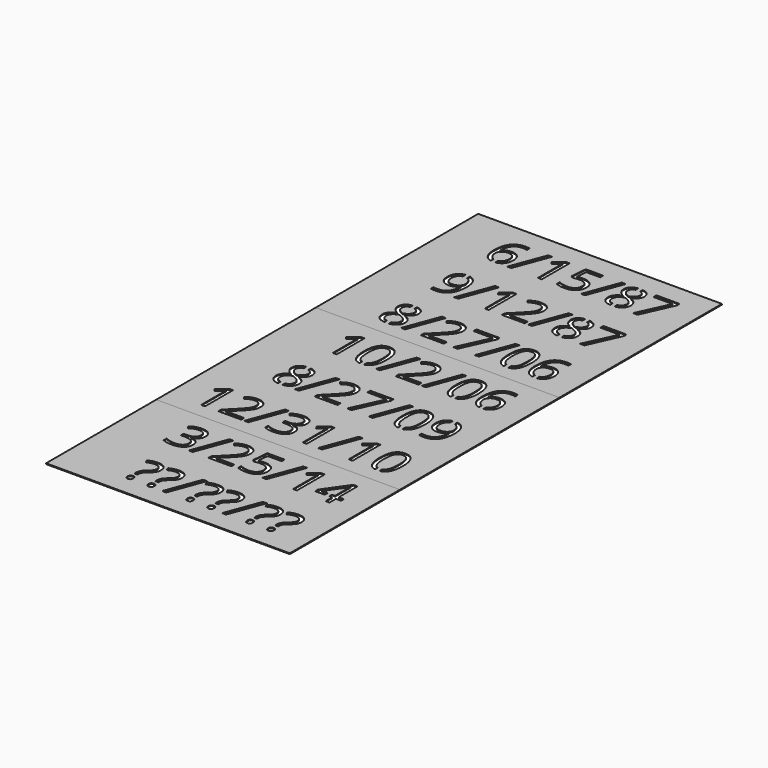
from build123d import *

# Parameters (mm, degrees)
F0_W     = 151.7277859016
F0_H     = 126.4366803746
F1_DEPTH = 0.508
F0_H_2   = 124.0870952606
F2_DEPTH = 0.508
F0_H_3   = 85.7449594557
F0_W_2   = 2.7546491474
F0_H_4   = 2.2408134275
F3_DEPTH = 0.508


with BuildPart() as f1:
    # F0 (on Top) → F1 (new body)
    with BuildSketch(Plane.XY):
        with Locations((63.5661068396, -28.6419243524)):
            Rectangle(F0_W, F0_H)
        with BuildLine():
            add(Edge.make_bspline(
                [(24.5445030092, -82.9433292213), (23.8799650872, -82.9433292213), (23.2740910724, -82.8875375825)],
                knots=[0, 0, 0, 0.1914867343, 0.1914867343, 0.1914867343], degree=2))
            add(Edge.make_bspline(
                [(23.2740910724, -82.8875375825), (20.7159129299, -82.6519688875), (19.2035811745, -81.4217599342)],
                knots=[0.1914867343, 0.1914867343, 0.1914867343, 1, 1, 1], degree=2))
            add(Edge.make_bspline(
                [(19.2035811745, -81.4217599342), (17.3330716609, -79.9001906471), (17.3330716609, -77.1086688348)],
                knots=[0, 0, 0, 1, 1, 1], degree=2))
            add(Edge.make_bspline(
                [(17.3330716609, -77.1086688348), (17.3330716609, -73.3866397518), (21.8716683488, -71.3072408508)],
                knots=[0, 0, 0, 1, 1, 1], degree=2))
            add(Edge.make_bspline(
                [(21.8716683488, -71.3072408508), (19.8255018504, -70.1536017345), (18.9353482113, -68.8100631752)],
                knots=[0, 0, 0, 1, 1, 1], degree=2))
            add(Edge.make_bspline(
                [(18.9353482113, -68.8100631752), (18.0451945722, -67.4665246159), (18.0451945722, -65.8049044896)],
                knots=[0, 0, 0, 1, 1, 1], degree=2))
            add(Edge.make_bspline(
                [(18.0451945722, -65.8049044896), (18.0451945722, -63.4454039101), (19.7875219618, -62.0448955179)],
                knots=[0, 0, 0, 1, 1, 1], degree=2))
            add(Edge.make_bspline(
                [(19.7875219618, -62.0448955179), (21.1170780871, -60.9761787415), (23.1349961832, -60.7229912076)],
                knots=[0, 0, 0, 0.7630920189, 0.7630920189, 0.7630920189], degree=2))
            add(Edge.make_bspline(
                [(23.1349961832, -60.7229912076), (23.7614748914, -60.6443871257), (24.4543007738, -60.6443871257)],
                knots=[0.7630920189, 0.7630920189, 0.7630920189, 1, 1, 1], degree=2))
            add(Edge.make_bspline(
                [(24.4543007738, -60.6443871257), (25.2121574841, -60.6443871257), (25.8896453306, -60.7343568942)],
                knots=[0, 0, 0, 0.2554132265, 0.2554132265, 0.2554132265], degree=2))
            add(Edge.make_bspline(
                [(25.8896453306, -60.7343568942), (27.864674175, -60.9966389247), (29.1566857314, -62.0235318306)],
                knots=[0.2554132265, 0.2554132265, 0.2554132265, 1, 1, 1], degree=2))
            add(Edge.make_bspline(
                [(29.1566857314, -62.0235318306), (30.8918918919, -63.4026765355), (30.8918918919, -65.833389406)],
                knots=[0, 0, 0, 1, 1, 1], degree=2))
            add(Edge.make_bspline(
                [(30.8918918919, -65.833389406), (30.8918918919, -67.4380396995), (29.8996673022, -68.7578408284)],
                knots=[0, 0, 0, 1, 1, 1], degree=2))
            add(Edge.make_bspline(
                [(29.8996673022, -68.7578408284), (28.9074427124, -70.0776419573), (26.7235991178, -71.1600687825)],
                knots=[0, 0, 0, 1, 1, 1], degree=2))
            add(Edge.make_bspline(
                [(26.7235991178, -71.1600687825), (29.3632013756, -72.4229000785), (30.4764868603, -73.8091660125)],
                knots=[0, 0, 0, 1, 1, 1], degree=2))
            add(Edge.make_bspline(
                [(30.4764868603, -73.8091660125), (31.589772345, -75.1954319465), (31.589772345, -77.0232140855)],
                knots=[0, 0, 0, 1, 1, 1], degree=2))
            add(Edge.make_bspline(
                [(31.589772345, -77.0232140855), (31.589772345, -79.7197861762), (29.7050203731, -81.3315576988)],
                knots=[0, 0, 0, 1, 1, 1], degree=2))
            add(Edge.make_bspline(
                [(29.7050203731, -81.3315576988), (28.2700445863, -82.5586969422), (26.0287402198, -82.8515407835)],
                knots=[0, 0, 0, 0.7613605441, 0.7613605441, 0.7613605441], degree=2))
            add(Edge.make_bspline(
                [(26.0287402198, -82.8515407835), (25.32622988, -82.9433292213), (24.5445030092, -82.9433292213)],
                knots=[0.7613605441, 0.7613605441, 0.7613605441, 1, 1, 1], degree=2))
        make_face(mode=Mode.SUBTRACT)
        Polygon((41.5452506448, -60.9529737206), (44.0044484318, -60.9529737206), (35.9194796456, -82.6442375986), (33.4602818586, -82.6442375986), align=None, mode=Mode.SUBTRACT)
        with BuildLine():
            Line((60.0604463385, -80.3606967964), (60.0604463385, -82.6442375986))
            Line((60.0604463385, -82.6442375986), (45.8037456544, -82.6442375986))
            Line((45.8037456544, -82.6442375986), (45.8037456544, -80.5221113229))
            Line((45.8037456544, -80.5221113229), (51.5149714029, -74.7824006579))
            add(Edge.make_bspline(
                [(51.5149714029, -74.7824006579), (54.1260887443, -72.138050914), (54.9568988075, -71.0105229711)],
                knots=[0, 0, 0, 1, 1, 1], degree=2))
            add(Edge.make_bspline(
                [(54.9568988075, -71.0105229711), (55.7877088707, -69.8829950282), (56.2031139023, -68.8148106613)],
                knots=[0, 0, 0, 1, 1, 1], degree=2))
            add(Edge.make_bspline(
                [(56.2031139023, -68.8148106613), (56.6185189339, -67.7466262943), (56.6185189339, -66.5170274008)],
                knots=[0, 0, 0, 1, 1, 1], degree=2))
            add(Edge.make_bspline(
                [(56.6185189339, -66.5170274008), (56.6185189339, -64.7794474973), (55.5645770252, -63.7634854772)],
                knots=[0, 0, 0, 1, 1, 1], degree=2))
            add(Edge.make_bspline(
                [(55.5645770252, -63.7634854772), (54.5106351164, -62.7475234571), (52.6401256028, -62.7475234571)],
                knots=[0, 0, 0, 1, 1, 1], degree=2))
            add(Edge.make_bspline(
                [(52.6401256028, -62.7475234571), (51.2918395574, -62.7475234571), (50.0812306082, -63.1937871481)],
                knots=[0, 0, 0, 1, 1, 1], degree=2))
            add(Edge.make_bspline(
                [(50.0812306082, -63.1937871481), (48.870621659, -63.6400508392), (47.3894060035, -64.8126798998)],
                knots=[0, 0, 0, 1, 1, 1], degree=2))
            Line((47.3894060035, -64.8126798998), (46.0838473328, -63.1368173152))
            add(Edge.make_bspline(
                [(46.0838473328, -63.1368173152), (49.0795110463, -60.6443871257), (52.6116406863, -60.6443871257)],
                knots=[0, 0, 0, 1, 1, 1], degree=2))
            add(Edge.make_bspline(
                [(52.6116406863, -60.6443871257), (55.6690217188, -60.6443871257), (57.4042278793, -62.2086837875)],
                knots=[0, 0, 0, 1, 1, 1], degree=2))
            add(Edge.make_bspline(
                [(57.4042278793, -62.2086837875), (59.1394340398, -63.7729804493), (59.1394340398, -66.4125827072)],
                knots=[0, 0, 0, 1, 1, 1], degree=2))
            add(Edge.make_bspline(
                [(59.1394340398, -66.4125827072), (59.1394340398, -68.4777391499), (57.9810474375, -70.4954207319)],
                knots=[0, 0, 0, 1, 1, 1], degree=2))
            add(Edge.make_bspline(
                [(57.9810474375, -70.4954207319), (56.8226608351, -72.5131023139), (53.6513401368, -75.5989682629)],
                knots=[0, 0, 0, 1, 1, 1], degree=2))
            Line((53.6513401368, -75.5989682629), (48.9038540615, -80.2420096445))
            Line((48.9038540615, -80.2420096445), (48.9038540615, -80.3606967964))
            Line((48.9038540615, -80.3606967964), (60.0604463385, -80.3606967964))
        make_face(mode=Mode.SUBTRACT)
        with BuildLine():
            add(Edge.make_bspline(
                [(19.2534297783, -21.2806063325), (20.7691418436, -19.7116446589), (23.0512460694, -19.39968802)],
                knots=[0, 0, 0, 0.8011700068, 0.8011700068, 0.8011700068], degree=2))
            add(Edge.make_bspline(
                [(23.0512460694, -19.39968802), (23.6176062225, -19.3222683264), (24.2311689283, -19.3222683264)],
                knots=[0.8011700068, 0.8011700068, 0.8011700068, 1, 1, 1], degree=2))
            add(Edge.make_bspline(
                [(24.2311689283, -19.3222683264), (25.0574379564, -19.3222683264), (25.8058952168, -19.480540773)],
                knots=[0, 0, 0, 0.3734838764, 0.3734838764, 0.3734838764], degree=2))
            add(Edge.make_bspline(
                [(25.8058952168, -19.480540773), (27.0614261009, -19.7460414975), (28.0979963366, -20.4569174984)],
                knots=[0.3734838764, 0.3734838764, 0.3734838764, 1, 1, 1], degree=2))
            add(Edge.make_bspline(
                [(28.0979963366, -20.4569174984), (29.7524952338, -21.5915666704), (30.6426488729, -23.7635415498)],
                knots=[0, 0, 0, 1, 1, 1], degree=2))
            add(Edge.make_bspline(
                [(30.6426488729, -23.7635415498), (31.5328025121, -25.9355164293), (31.5328025121, -28.8884527681)],
                knots=[0, 0, 0, 1, 1, 1], degree=2))
            add(Edge.make_bspline(
                [(31.5328025121, -28.8884527681), (31.5328025121, -41.621210422), (21.6817689058, -41.621210422)],
                knots=[0, 0, 0, 1, 1, 1], degree=2))
            add(Edge.make_bspline(
                [(21.6817689058, -41.621210422), (19.9584314605, -41.621210422), (18.9519644125, -41.3221187993)],
                knots=[0, 0, 0, 1, 1, 1], degree=2))
            Line((18.9519644125, -41.3221187993), (18.9519644125, -39.1999925236))
            add(Edge.make_bspline(
                [(18.9519644125, -39.1999925236), (20.1388359314, -39.5845388957), (21.6485365033, -39.5845388957)],
                knots=[0, 0, 0, 1, 1, 1], degree=2))
            add(Edge.make_bspline(
                [(21.6485365033, -39.5845388957), (25.2091510598, -39.5845388957), (27.0274382266, -37.3817053568)],
                knots=[0, 0, 0, 1, 1, 1], degree=2))
            add(Edge.make_bspline(
                [(27.0274382266, -37.3817053568), (28.8457253934, -35.1788718179), (29.00713992, -30.6260326717)],
                knots=[0, 0, 0, 1, 1, 1], degree=2))
            Line((29.00713992, -30.6260326717), (28.8314829352, -30.6260326717))
            add(Edge.make_bspline(
                [(28.8314829352, -30.6260326717), (28.0149153303, -31.8556315652), (26.6642555418, -32.5012896714)],
                knots=[0, 0, 0, 1, 1, 1], degree=2))
            add(Edge.make_bspline(
                [(26.6642555418, -32.5012896714), (25.3135957534, -33.1469477777), (23.6234907106, -33.1469477777)],
                knots=[0, 0, 0, 1, 1, 1], degree=2))
            add(Edge.make_bspline(
                [(23.6234907106, -33.1469477777), (20.746514149, -33.1469477777), (19.0540353632, -31.4259840754)],
                knots=[0, 0, 0, 1, 1, 1], degree=2))
            add(Edge.make_bspline(
                [(19.0540353632, -31.4259840754), (17.3615565773, -29.7050203731), (17.3615565773, -26.6191544241)],
                knots=[0, 0, 0, 1, 1, 1], degree=2))
            add(Edge.make_bspline(
                [(17.3615565773, -26.6191544241), (17.3615565773, -23.2389443385), (19.2534297783, -21.2806063325)],
                knots=[0, 0, 0, 1, 1, 1], degree=2))
        make_face(mode=Mode.SUBTRACT)
        with BuildLine():
            add(Edge.make_bspline(
                [(24.8388471459, -0.2990916227), (24.0678679787, -0.2990916227), (23.3699921519, -0.1663349604)],
                knots=[0, 0, 0, 0.2290512722, 0.2290512722, 0.2290512722], degree=2))
            add(Edge.make_bspline(
                [(23.3699921519, -0.1663349604), (21.0210574537, 0.2805020248), (19.5002990542, 2.2313184554)],
                knots=[0.2290512722, 0.2290512722, 0.2290512722, 1, 1, 1], degree=2))
            add(Edge.make_bspline(
                [(19.5002990542, 2.2313184554), (17.52771859, 4.7617285335), (17.52771859, 9.271840305)],
                knots=[0, 0, 0, 1, 1, 1], degree=2))
            add(Edge.make_bspline(
                [(17.52771859, 9.271840305), (17.52771859, 15.6667040484), (20.0130275504, 18.8332772607)],
                knots=[0, 0, 0, 1, 1, 1], degree=2))
            add(Edge.make_bspline(
                [(20.0130275504, 18.8332772607), (22.4983365108, 21.9998504729), (27.364509738, 21.9998504729)],
                knots=[0, 0, 0, 1, 1, 1], degree=2))
            add(Edge.make_bspline(
                [(27.364509738, 21.9998504729), (29.0403723225, 21.9998504729), (30.0041119958, 21.7197487944)],
                knots=[0, 0, 0, 1, 1, 1], degree=2))
            Line((30.0041119958, 21.7197487944), (30.0041119958, 19.5976225188))
            add(Edge.make_bspline(
                [(30.0041119958, 19.5976225188), (28.8599678517, 19.9679264327), (27.3929946544, 19.9679264327)],
                knots=[0, 0, 0, 1, 1, 1], degree=2))
            add(Edge.make_bspline(
                [(27.3929946544, 19.9679264327), (23.9035923891, 19.9679264327), (22.0639415349, 17.7959515532)],
                knots=[0, 0, 0, 1, 1, 1], degree=2))
            add(Edge.make_bspline(
                [(22.0639415349, 17.7959515532), (20.2242906807, 15.6239766738), (20.0486336959, 10.9619453478)],
                knots=[0, 0, 0, 1, 1, 1], degree=2))
            Line((20.0486336959, 10.9619453478), (20.2242906807, 10.9619453478))
            add(Edge.make_bspline(
                [(20.2242906807, 10.9619453478), (21.8574258906, 13.5160928563), (25.3895555306, 13.5160928563)],
                knots=[0, 0, 0, 1, 1, 1], degree=2))
            add(Edge.make_bspline(
                [(25.3895555306, 13.5160928563), (28.314006953, 13.5160928563), (29.9969907667, 11.7500280363)],
                knots=[0, 0, 0, 1, 1, 1], degree=2))
            add(Edge.make_bspline(
                [(29.9969907667, 11.7500280363), (31.6799745804, 9.9839632163), (31.6799745804, 6.9598145864)],
                knots=[0, 0, 0, 1, 1, 1], degree=2))
            add(Edge.make_bspline(
                [(31.6799745804, 6.9598145864), (31.6799745804, 3.5748570147), (29.8332024971, 1.637882696)],
                knots=[0, 0, 0, 1, 1, 1], degree=2))
            add(Edge.make_bspline(
                [(29.8332024971, 1.637882696), (28.3810605434, 0.1148135003), (26.1246412992, -0.2106457155)],
                knots=[0, 0, 0, 0.7863135721, 0.7863135721, 0.7863135721], degree=2))
            add(Edge.make_bspline(
                [(26.1246412992, -0.2106457155), (25.5114429708, -0.2990916227), (24.8388471459, -0.2990916227)],
                knots=[0.7863135721, 0.7863135721, 0.7863135721, 1, 1, 1], degree=2))
        make_face(mode=Mode.SUBTRACT)
        Polygon((41.5452506448, -19.6308549213), (44.0044484318, -19.6308549213), (35.9194796456, -41.3221187993), (33.4602818586, -41.3221187993), align=None, mode=Mode.SUBTRACT)
        with BuildLine():
            Line((54.923666405, -19.6308549213), (54.923666405, -41.3221187993))
            Line((54.923666405, -41.3221187993), (52.5214384509, -41.3221187993))
            Line((52.5214384509, -41.3221187993), (52.5214384509, -25.8643041382))
            add(Edge.make_bspline(
                [(52.5214384509, -25.8643041382), (52.5214384509, -23.9320773055), (52.6401256028, -22.2134873463)],
                knots=[0, 0, 0, 1, 1, 1], degree=2))
            add(Edge.make_bspline(
                [(52.6401256028, -22.2134873463), (52.3315390079, -22.5268214272), (51.9446188928, -22.8662666816)],
                knots=[0, 0, 0, 1, 1, 1], degree=2))
            add(Edge.make_bspline(
                [(51.9446188928, -22.8662666816), (51.5576987776, -23.205711936), (48.4148629958, -25.7598594445)],
                knots=[0, 0, 0, 1, 1, 1], degree=2))
            Line((48.4148629958, -25.7598594445), (47.1093043251, -24.0697544017))
            Line((47.1093043251, -24.0697544017), (52.8490149901, -19.6308549213))
            Line((52.8490149901, -19.6308549213), (54.923666405, -19.6308549213))
        make_face(mode=Mode.SUBTRACT)
        Polygon((41.5452506448, 21.691263878), (44.0044484318, 21.691263878), (35.9194796456, 0), (33.4602818586, 0), align=None, mode=Mode.SUBTRACT)
        with BuildLine():
            Line((54.923666405, 21.691263878), (54.923666405, 0))
            Line((54.923666405, 0), (52.5214384509, 0))
            Line((52.5214384509, 0), (52.5214384509, 15.4578146611))
            add(Edge.make_bspline(
                [(52.5214384509, 15.4578146611), (52.5214384509, 17.3900414938), (52.6401256028, 19.108631453)],
                knots=[0, 0, 0, 1, 1, 1], degree=2))
            add(Edge.make_bspline(
                [(52.6401256028, 19.108631453), (52.3315390079, 18.7952973721), (51.9446188928, 18.4558521177)],
                knots=[0, 0, 0, 1, 1, 1], degree=2))
            add(Edge.make_bspline(
                [(51.9446188928, 18.4558521177), (51.5576987776, 18.1164068633), (48.4148629958, 15.5622593548)],
                knots=[0, 0, 0, 1, 1, 1], degree=2))
            Line((48.4148629958, 15.5622593548), (47.1093043251, 17.2523643976))
            Line((47.1093043251, 17.2523643976), (52.8490149901, 21.691263878))
            Line((52.8490149901, 21.691263878), (54.923666405, 21.691263878))
        make_face(mode=Mode.SUBTRACT)
        Polygon((68.6486486486, -82.6442375986), (65.9188441554, -82.6442375986), (74.9058352959, -63.2222720646), (63.0845949684, -63.2222720646), (63.0845949684, -60.9529737206), (77.5169526373, -60.9529737206), (77.5169526373, -62.9279279279), align=None, mode=Mode.SUBTRACT)
        Polygon((87.4439460207, -60.9529737206), (89.9031438077, -60.9529737206), (81.8181750215, -82.6442375986), (79.3589772345, -82.6442375986), align=None, mode=Mode.SUBTRACT)
        with BuildLine():
            add(Edge.make_bspline(
                [(98.8806399761, -82.9433292213), (98.1965363244, -82.9433292213), (97.5764067844, -82.8347093468)],
                knots=[0, 0, 0, 0.1955197896, 0.1955197896, 0.1955197896], degree=2))
            add(Edge.make_bspline(
                [(97.5764067844, -82.8347093468), (95.0248392731, -82.3877850755), (93.5563343426, -80.1019588053)],
                knots=[0.1955197896, 0.1955197896, 0.1955197896, 1, 1, 1], degree=2))
            add(Edge.make_bspline(
                [(93.5563343426, -80.1019588053), (91.7309259467, -77.2605883892), (91.7309259467, -71.7677470001)],
                knots=[0, 0, 0, 1, 1, 1], degree=2))
            add(Edge.make_bspline(
                [(91.7309259467, -71.7677470001), (91.7309259467, -66.1039961123), (93.4969907667, -63.3575754177)],
                knots=[0, 0, 0, 1, 1, 1], degree=2))
            add(Edge.make_bspline(
                [(93.4969907667, -63.3575754177), (95.2630555867, -60.6111547232), (98.8806399761, -60.6111547232)],
                knots=[0, 0, 0, 1, 1, 1], degree=2))
            add(Edge.make_bspline(
                [(98.8806399761, -60.6111547232), (102.4127696161, -60.6111547232), (104.2452992411, -63.4762625696)],
                knots=[0, 0, 0, 1, 1, 1], degree=2))
            add(Edge.make_bspline(
                [(104.2452992411, -63.4762625696), (106.0778288662, -66.3413704161), (106.0778288662, -71.7677470001)],
                knots=[0, 0, 0, 1, 1, 1], degree=2))
            add(Edge.make_bspline(
                [(106.0778288662, -71.7677470001), (106.0778288662, -77.3935179993), (104.3046428171, -80.1684236103)],
                knots=[0, 0, 0, 1, 1, 1], degree=2))
            add(Edge.make_bspline(
                [(104.3046428171, -80.1684236103), (102.9037921932, -82.3606516951), (100.3310559317, -82.8209779967)],
                knots=[0, 0, 0, 0.7900189744, 0.7900189744, 0.7900189744], degree=2))
            add(Edge.make_bspline(
                [(100.3310559317, -82.8209779967), (99.6472422305, -82.9433292213), (98.8806399761, -82.9433292213)],
                knots=[0.7900189744, 0.7900189744, 0.7900189744, 1, 1, 1], degree=2))
        make_face(mode=Mode.SUBTRACT)
        with BuildLine():
            add(Edge.make_bspline(
                [(116.6362378976, -82.9433292213), (115.9879006736, -82.9433292213), (115.3912590817, -82.8494492489)],
                knots=[0, 0, 0, 0.1926154069, 0.1926154069, 0.1926154069], degree=2))
            add(Edge.make_bspline(
                [(115.3912590817, -82.8494492489), (112.8903208816, -82.4559332546), (111.297689806, -80.4129191432)],
                knots=[0.1926154069, 0.1926154069, 0.1926154069, 1, 1, 1], degree=2))
            add(Edge.make_bspline(
                [(111.297689806, -80.4129191432), (109.3251093417, -77.8825090651), (109.3251093417, -73.3723972936)],
                knots=[0, 0, 0, 1, 1, 1], degree=2))
            add(Edge.make_bspline(
                [(109.3251093417, -73.3723972936), (109.3251093417, -66.9775335501), (111.8104183021, -63.8109603379)],
                knots=[0, 0, 0, 1, 1, 1], degree=2))
            add(Edge.make_bspline(
                [(111.8104183021, -63.8109603379), (114.2957272625, -60.6443871257), (119.1619004897, -60.6443871257)],
                knots=[0, 0, 0, 1, 1, 1], degree=2))
            add(Edge.make_bspline(
                [(119.1619004897, -60.6443871257), (120.8377630743, -60.6443871257), (121.8015027476, -60.9244888042)],
                knots=[0, 0, 0, 1, 1, 1], degree=2))
            Line((121.8015027476, -60.9244888042), (121.8015027476, -63.0466150798))
            add(Edge.make_bspline(
                [(121.8015027476, -63.0466150798), (120.6573586034, -62.6763111659), (119.1903854062, -62.6763111659)],
                knots=[0, 0, 0, 1, 1, 1], degree=2))
            add(Edge.make_bspline(
                [(119.1903854062, -62.6763111659), (115.7009831408, -62.6763111659), (113.8613322866, -64.8482860454)],
                knots=[0, 0, 0, 1, 1, 1], degree=2))
            add(Edge.make_bspline(
                [(113.8613322866, -64.8482860454), (112.0216814325, -67.0202609248), (111.8460244477, -71.6822922508)],
                knots=[0, 0, 0, 1, 1, 1], degree=2))
            Line((111.8460244477, -71.6822922508), (112.0216814325, -71.6822922508))
            add(Edge.make_bspline(
                [(112.0216814325, -71.6822922508), (113.6548166424, -69.1281447423), (117.1869462824, -69.1281447423)],
                knots=[0, 0, 0, 1, 1, 1], degree=2))
            add(Edge.make_bspline(
                [(117.1869462824, -69.1281447423), (120.1113977048, -69.1281447423), (121.7943815184, -70.8942095623)],
                knots=[0, 0, 0, 1, 1, 1], degree=2))
            add(Edge.make_bspline(
                [(121.7943815184, -70.8942095623), (123.4773653321, -72.6602743823), (123.4773653321, -75.6844230122)],
                knots=[0, 0, 0, 1, 1, 1], degree=2))
            add(Edge.make_bspline(
                [(123.4773653321, -75.6844230122), (123.4773653321, -79.0693805839), (121.6305932489, -81.0063549026)],
                knots=[0, 0, 0, 1, 1, 1], degree=2))
            add(Edge.make_bspline(
                [(121.6305932489, -81.0063549026), (120.2511386429, -82.4531864688), (118.1459082291, -82.8193007737)],
                knots=[0, 0, 0, 0.7469544393, 0.7469544393, 0.7469544393], degree=2))
            add(Edge.make_bspline(
                [(118.1459082291, -82.8193007737), (117.4327198705, -82.9433292213), (116.6362378976, -82.9433292213)],
                knots=[0.7469544393, 0.7469544393, 0.7469544393, 1, 1, 1], degree=2))
        make_face(mode=Mode.SUBTRACT)
        with BuildLine():
            Line((77.4314978879, -39.0385779971), (77.4314978879, -41.3221187993))
            Line((77.4314978879, -41.3221187993), (63.1747972038, -41.3221187993))
            Line((63.1747972038, -41.3221187993), (63.1747972038, -39.1999925236))
            Line((63.1747972038, -39.1999925236), (68.8860229524, -33.4602818586))
            add(Edge.make_bspline(
                [(68.8860229524, -33.4602818586), (71.4971402938, -30.8159321147), (72.327950357, -29.6884041718)],
                knots=[0, 0, 0, 1, 1, 1], degree=2))
            add(Edge.make_bspline(
                [(72.327950357, -29.6884041718), (73.1587604202, -28.5608762289), (73.5741654518, -27.492691862)],
                knots=[0, 0, 0, 1, 1, 1], degree=2))
            add(Edge.make_bspline(
                [(73.5741654518, -27.492691862), (73.9895704833, -26.424507495), (73.9895704833, -25.1949086015)],
                knots=[0, 0, 0, 1, 1, 1], degree=2))
            add(Edge.make_bspline(
                [(73.9895704833, -25.1949086015), (73.9895704833, -23.457328698), (72.9356285746, -22.4413666779)],
                knots=[0, 0, 0, 1, 1, 1], degree=2))
            add(Edge.make_bspline(
                [(72.9356285746, -22.4413666779), (71.8816866659, -21.4254046578), (70.0111771523, -21.4254046578)],
                knots=[0, 0, 0, 1, 1, 1], degree=2))
            add(Edge.make_bspline(
                [(70.0111771523, -21.4254046578), (68.6628911069, -21.4254046578), (67.4522821577, -21.8716683488)],
                knots=[0, 0, 0, 1, 1, 1], degree=2))
            add(Edge.make_bspline(
                [(67.4522821577, -21.8716683488), (66.2416732085, -22.3179320399), (64.760457553, -23.4905611005)],
                knots=[0, 0, 0, 1, 1, 1], degree=2))
            Line((64.760457553, -23.4905611005), (63.4548988823, -21.8146985159))
            add(Edge.make_bspline(
                [(63.4548988823, -21.8146985159), (66.4505625958, -19.3222683264), (69.9826922358, -19.3222683264)],
                knots=[0, 0, 0, 1, 1, 1], degree=2))
            add(Edge.make_bspline(
                [(69.9826922358, -19.3222683264), (73.0400732683, -19.3222683264), (74.7752794288, -20.8865649882)],
                knots=[0, 0, 0, 1, 1, 1], degree=2))
            add(Edge.make_bspline(
                [(74.7752794288, -20.8865649882), (76.5104855893, -22.45086165), (76.5104855893, -25.0904639079)],
                knots=[0, 0, 0, 1, 1, 1], degree=2))
            add(Edge.make_bspline(
                [(76.5104855893, -25.0904639079), (76.5104855893, -27.1556203506), (75.352098987, -29.1733019326)],
                knots=[0, 0, 0, 1, 1, 1], degree=2))
            add(Edge.make_bspline(
                [(75.352098987, -29.1733019326), (74.1937123846, -31.1909835146), (71.0223916863, -34.2768494636)],
                knots=[0, 0, 0, 1, 1, 1], degree=2))
            Line((71.0223916863, -34.2768494636), (66.274905611, -38.9198908452))
            Line((66.274905611, -38.9198908452), (66.274905611, -39.0385779971))
            Line((66.274905611, -39.0385779971), (77.4314978879, -39.0385779971))
        make_face(mode=Mode.SUBTRACT)
        Polygon((87.4439460207, -19.6308549213), (89.9031438077, -19.6308549213), (81.8181750215, -41.3221187993), (79.3589772345, -41.3221187993), align=None, mode=Mode.SUBTRACT)
        with BuildLine():
            add(Edge.make_bspline(
                [(98.9708422115, -41.621210422), (98.316182622, -41.621210422), (97.7184558287, -41.5670651365)],
                knots=[0, 0, 0, 0.1886402908, 0.1886402908, 0.1886402908], degree=2))
            add(Edge.make_bspline(
                [(97.7184558287, -41.5670651365), (95.1475764318, -41.3341811492), (93.6299203768, -40.0996411349)],
                knots=[0.1886402908, 0.1886402908, 0.1886402908, 1, 1, 1], degree=2))
            add(Edge.make_bspline(
                [(93.6299203768, -40.0996411349), (91.7594108631, -38.5780718478), (91.7594108631, -35.7865500355)],
                knots=[0, 0, 0, 1, 1, 1], degree=2))
            add(Edge.make_bspline(
                [(91.7594108631, -35.7865500355), (91.7594108631, -32.0645209525), (96.2980075511, -29.9851220515)],
                knots=[0, 0, 0, 1, 1, 1], degree=2))
            add(Edge.make_bspline(
                [(96.2980075511, -29.9851220515), (94.2518410527, -28.8314829352), (93.3616874136, -27.4879443759)],
                knots=[0, 0, 0, 1, 1, 1], degree=2))
            add(Edge.make_bspline(
                [(93.3616874136, -27.4879443759), (92.4715337744, -26.1444058166), (92.4715337744, -24.4827856903)],
                knots=[0, 0, 0, 1, 1, 1], degree=2))
            add(Edge.make_bspline(
                [(92.4715337744, -24.4827856903), (92.4715337744, -22.1232851108), (94.2138611641, -20.7227767186)],
                knots=[0, 0, 0, 1, 1, 1], degree=2))
            add(Edge.make_bspline(
                [(94.2138611641, -20.7227767186), (95.5493510675, -19.649290284), (97.5793609396, -19.3986287119)],
                knots=[0, 0, 0, 0.7664976808, 0.7664976808, 0.7664976808], degree=2))
            add(Edge.make_bspline(
                [(97.5793609396, -19.3986287119), (98.1977737866, -19.3222683264), (98.8806399761, -19.3222683264)],
                knots=[0.7664976808, 0.7664976808, 0.7664976808, 1, 1, 1], degree=2))
            add(Edge.make_bspline(
                [(98.8806399761, -19.3222683264), (99.6485865968, -19.3222683264), (100.334010087, -19.4146497116)],
                knots=[0, 0, 0, 0.2588137329, 0.2588137329, 0.2588137329], degree=2))
            add(Edge.make_bspline(
                [(100.334010087, -19.4146497116), (102.296913957, -19.6792099157), (103.5830249336, -20.7014130313)],
                knots=[0.2588137329, 0.2588137329, 0.2588137329, 1, 1, 1], degree=2))
            add(Edge.make_bspline(
                [(103.5830249336, -20.7014130313), (105.3182310942, -22.0805577362), (105.3182310942, -24.5112706067)],
                knots=[0, 0, 0, 1, 1, 1], degree=2))
            add(Edge.make_bspline(
                [(105.3182310942, -24.5112706067), (105.3182310942, -26.1159209002), (104.3260065044, -27.4357220291)],
                knots=[0, 0, 0, 1, 1, 1], degree=2))
            add(Edge.make_bspline(
                [(104.3260065044, -27.4357220291), (103.3337819147, -28.755523158), (101.1499383201, -29.8379499832)],
                knots=[0, 0, 0, 1, 1, 1], degree=2))
            add(Edge.make_bspline(
                [(101.1499383201, -29.8379499832), (103.7895405779, -31.1007812792), (104.9028260626, -32.4870472132)],
                knots=[0, 0, 0, 1, 1, 1], degree=2))
            add(Edge.make_bspline(
                [(104.9028260626, -32.4870472132), (106.0161115472, -33.8733131472), (106.0161115472, -35.7010952862)],
                knots=[0, 0, 0, 1, 1, 1], degree=2))
            add(Edge.make_bspline(
                [(106.0161115472, -35.7010952862), (106.0161115472, -38.3976673769), (104.1313595753, -40.0094388995)],
                knots=[0, 0, 0, 1, 1, 1], degree=2))
            add(Edge.make_bspline(
                [(104.1313595753, -40.0094388995), (102.7021583212, -41.231639972), (100.4731049761, -41.5270499697)],
                knots=[0, 0, 0, 0.7582967284, 0.7582967284, 0.7582967284], degree=2))
            add(Edge.make_bspline(
                [(100.4731049761, -41.5270499697), (99.7626054237, -41.621210422), (98.9708422115, -41.621210422)],
                knots=[0.7582967284, 0.7582967284, 0.7582967284, 1, 1, 1], degree=2))
        make_face(mode=Mode.SUBTRACT)
        with BuildLine():
            add(Edge.make_bspline(
                [(66.5550072894, 12.9084146387), (68.2593547905, 13.2502336361), (69.9542073194, 13.2502336361)],
                knots=[0, 0, 0, 1, 1, 1], degree=2))
            add(Edge.make_bspline(
                [(69.9542073194, 13.2502336361), (73.3818922657, 13.2502336361), (75.3473515009, 11.5506336212)],
                knots=[0, 0, 0, 1, 1, 1], degree=2))
            add(Edge.make_bspline(
                [(75.3473515009, 11.5506336212), (77.312810736, 9.8510336062), (77.312810736, 6.8980972674)],
                knots=[0, 0, 0, 1, 1, 1], degree=2))
            add(Edge.make_bspline(
                [(77.312810736, 6.8980972674), (77.312810736, 3.53212964), (75.1693207731, 1.6165190086)],
                knots=[0, 0, 0, 1, 1, 1], degree=2))
            add(Edge.make_bspline(
                [(75.1693207731, 1.6165190086), (73.0258308101, -0.2990916227), (69.2563268663, -0.2990916227)],
                knots=[0, 0, 0, 1, 1, 1], degree=2))
            add(Edge.make_bspline(
                [(69.2563268663, -0.2990916227), (65.5912676162, -0.2990916227), (63.6637882696, 0.8735374379)],
                knots=[0, 0, 0, 1, 1, 1], degree=2))
            Line((63.6637882696, 0.8735374379), (63.6637882696, 3.2472804755))
            add(Edge.make_bspline(
                [(63.6637882696, 3.2472804755), (64.698740234, 2.582632425), (66.2416732085, 2.2028335389)],
                knots=[0, 0, 0, 1, 1, 1], degree=2))
            add(Edge.make_bspline(
                [(66.2416732085, 2.2028335389), (67.7846061829, 1.8230346529), (69.2848117827, 1.8230346529)],
                knots=[0, 0, 0, 1, 1, 1], degree=2))
            add(Edge.make_bspline(
                [(69.2848117827, 1.8230346529), (71.8959291241, 1.8230346529), (73.3415386341, 3.0550072894)],
                knots=[0, 0, 0, 1, 1, 1], degree=2))
            add(Edge.make_bspline(
                [(73.3415386341, 3.0550072894), (74.787148144, 4.286979926), (74.787148144, 6.6179955889)],
                knots=[0, 0, 0, 1, 1, 1], degree=2))
            add(Edge.make_bspline(
                [(74.787148144, 6.6179955889), (74.787148144, 11.1565922769), (69.2278419498, 11.1565922769)],
                knots=[0, 0, 0, 1, 1, 1], degree=2))
            add(Edge.make_bspline(
                [(69.2278419498, 11.1565922769), (67.8178385855, 11.1565922769), (65.4583380061, 10.7245710441)],
                knots=[0, 0, 0, 1, 1, 1], degree=2))
            Line((65.4583380061, 10.7245710441), (64.1812642518, 11.541138649))
            Line((64.1812642518, 11.541138649), (64.9978318568, 21.691263878))
            Line((64.9978318568, 21.691263878), (75.7841202198, 21.691263878))
            Line((75.7841202198, 21.691263878), (75.7841202198, 19.421965534))
            Line((75.7841202198, 19.421965534), (67.1057156742, 19.421965534))
            Line((67.1057156742, 19.421965534), (66.5550072894, 12.9084146387))
        make_face(mode=Mode.SUBTRACT)
        Polygon((87.4439460207, 21.691263878), (89.9031438077, 21.691263878), (81.8181750215, 0), (79.3589772345, 0), align=None, mode=Mode.SUBTRACT)
        with BuildLine():
            add(Edge.make_bspline(
                [(98.9708422115, -0.2990916227), (98.2727327705, -0.2990916227), (97.6393641904, -0.2375205666)],
                knots=[0, 0, 0, 0.2011603742, 0.2011603742, 0.2011603742], degree=2))
            add(Edge.make_bspline(
                [(97.6393641904, -0.2375205666), (95.1241574968, 0.0069878244), (93.6299203768, 1.2224776644)],
                knots=[0.2011603742, 0.2011603742, 0.2011603742, 1, 1, 1], degree=2))
            add(Edge.make_bspline(
                [(93.6299203768, 1.2224776644), (91.7594108631, 2.7440469515), (91.7594108631, 5.5355687638)],
                knots=[0, 0, 0, 1, 1, 1], degree=2))
            add(Edge.make_bspline(
                [(91.7594108631, 5.5355687638), (91.7594108631, 9.2575978468), (96.2980075511, 11.3369967478)],
                knots=[0, 0, 0, 1, 1, 1], degree=2))
            add(Edge.make_bspline(
                [(96.2980075511, 11.3369967478), (94.2518410527, 12.4906358641), (93.3616874136, 13.8341744234)],
                knots=[0, 0, 0, 1, 1, 1], degree=2))
            add(Edge.make_bspline(
                [(93.3616874136, 13.8341744234), (92.4715337744, 15.1777129827), (92.4715337744, 16.839333109)],
                knots=[0, 0, 0, 1, 1, 1], degree=2))
            add(Edge.make_bspline(
                [(92.4715337744, 16.839333109), (92.4715337744, 19.1988336885), (94.2138611641, 20.5993420807)],
                knots=[0, 0, 0, 1, 1, 1], degree=2))
            add(Edge.make_bspline(
                [(94.2138611641, 20.5993420807), (95.5232476378, 21.6518461944), (97.5002693012, 21.9133768905)],
                knots=[0, 0, 0, 0.7515157493, 0.7515157493, 0.7515157493], degree=2))
            add(Edge.make_bspline(
                [(97.5002693012, 21.9133768905), (98.1539598556, 21.9998504729), (98.8806399761, 21.9998504729)],
                knots=[0.7515157493, 0.7515157493, 0.7515157493, 1, 1, 1], degree=2))
            add(Edge.make_bspline(
                [(98.8806399761, 21.9998504729), (99.6044323951, 21.9998504729), (100.2549184486, 21.9177868922)],
                knots=[0, 0, 0, 0.243932863, 0.243932863, 0.243932863], degree=2))
            add(Edge.make_bspline(
                [(100.2549184486, 21.9177868922), (102.2710925798, 21.6634317565), (103.5830249336, 20.620705768)],
                knots=[0.243932863, 0.243932863, 0.243932863, 1, 1, 1], degree=2))
            add(Edge.make_bspline(
                [(103.5830249336, 20.620705768), (105.3182310942, 19.2415610631), (105.3182310942, 16.8108481926)],
                knots=[0, 0, 0, 1, 1, 1], degree=2))
            add(Edge.make_bspline(
                [(105.3182310942, 16.8108481926), (105.3182310942, 15.2061978991), (104.3260065044, 13.8863967702)],
                knots=[0, 0, 0, 1, 1, 1], degree=2))
            add(Edge.make_bspline(
                [(104.3260065044, 13.8863967702), (103.3337819147, 12.5665956413), (101.1499383201, 11.4841688161)],
                knots=[0, 0, 0, 1, 1, 1], degree=2))
            add(Edge.make_bspline(
                [(101.1499383201, 11.4841688161), (103.7895405779, 10.2213375201), (104.9028260626, 8.8350715861)],
                knots=[0, 0, 0, 1, 1, 1], degree=2))
            add(Edge.make_bspline(
                [(104.9028260626, 8.8350715861), (106.0161115472, 7.4488056521), (106.0161115472, 5.6210235131)],
                knots=[0, 0, 0, 1, 1, 1], degree=2))
            add(Edge.make_bspline(
                [(106.0161115472, 5.6210235131), (106.0161115472, 2.9244514224), (104.1313595753, 1.3126798998)],
                knots=[0, 0, 0, 1, 1, 1], degree=2))
            add(Edge.make_bspline(
                [(104.1313595753, 1.3126798998), (102.6768829415, 0.0688642394), (100.3940133378, -0.2150899422)],
                knots=[0, 0, 0, 0.7717071824, 0.7717071824, 0.7717071824], degree=2))
            add(Edge.make_bspline(
                [(100.3940133378, -0.2150899422), (99.7186759225, -0.2990916227), (98.9708422115, -0.2990916227)],
                knots=[0.7717071824, 0.7717071824, 0.7717071824, 1, 1, 1], degree=2))
        make_face(mode=Mode.SUBTRACT)
        Polygon((114.5473440245, -41.3221187993), (111.8175395312, -41.3221187993), (120.8045306718, -21.9001532653), (108.9832903443, -21.9001532653), (108.9832903443, -19.6308549213), (123.4156480132, -19.6308549213), (123.4156480132, -21.6058091286), align=None, mode=Mode.SUBTRACT)
        Polygon((114.5473440245, 0), (111.8175395312, 0), (120.8045306718, 19.421965534), (108.9832903443, 19.421965534), (108.9832903443, 21.691263878), (123.4156480132, 21.691263878), (123.4156480132, 19.7163096707), align=None, mode=Mode.SUBTRACT)
        with BuildLine():
            add(Edge.make_bspline(
                [(24.4258158574, -62.6430787634), (23.7228789611, -62.6430787634), (23.1349961832, -62.7707275635)],
                knots=[0, 0, 0, 0.3786830641, 0.3786830641, 0.3786830641], degree=2))
            add(Edge.make_bspline(
                [(23.1349961832, -62.7707275635), (22.1704388506, -62.980164871), (21.5156068932, -63.5332324025)],
                knots=[0.3786830641, 0.3786830641, 0.3786830641, 1, 1, 1], degree=2))
            add(Edge.make_bspline(
                [(21.5156068932, -63.5332324025), (20.4616649845, -64.4233860416), (20.4616649845, -65.9093491832)],
                knots=[0, 0, 0, 1, 1, 1], degree=2))
            add(Edge.make_bspline(
                [(20.4616649845, -65.9093491832), (20.4616649845, -67.2718776868), (21.3375761654, -68.2522335614)],
                knots=[0, 0, 0, 1, 1, 1], degree=2))
            add(Edge.make_bspline(
                [(21.3375761654, -68.2522335614), (22.2134873463, -69.2325894359), (24.5729879257, -70.2105715674)],
                knots=[0, 0, 0, 1, 1, 1], degree=2))
            add(Edge.make_bspline(
                [(24.5729879257, -70.2105715674), (26.6951142013, -69.3227916713), (27.5781466113, -68.2973346791)],
                knots=[0, 0, 0, 1, 1, 1], degree=2))
            add(Edge.make_bspline(
                [(27.5781466113, -68.2973346791), (28.4611790213, -67.2718776868), (28.4611790213, -65.9093491832)],
                knots=[0, 0, 0, 1, 1, 1], degree=2))
            add(Edge.make_bspline(
                [(28.4611790213, -65.9093491832), (28.4611790213, -64.4091435834), (27.3858734253, -63.5261111734)],
                knots=[0, 0, 0, 1, 1, 1], degree=2))
            add(Edge.make_bspline(
                [(27.3858734253, -63.5261111734), (26.7703650731, -63.020660606), (25.8896453306, -62.8045315552)],
                knots=[0, 0, 0, 0.5724031889, 0.5724031889, 0.5724031889], degree=2))
            add(Edge.make_bspline(
                [(25.8896453306, -62.8045315552), (25.2317297902, -62.6430787634), (24.4258158574, -62.6430787634)],
                knots=[0.5724031889, 0.5724031889, 0.5724031889, 1, 1, 1], degree=2))
        make_face()
        with BuildLine():
            add(Edge.make_bspline(
                [(21.0052521401, -79.9452917648), (21.8853945714, -80.6531222422), (23.2740910724, -80.8572076717)],
                knots=[0, 0, 0, 0.7116747073, 0.7116747073, 0.7116747073], degree=2))
            add(Edge.make_bspline(
                [(23.2740910724, -80.8572076717), (23.8367025029, -80.9398900976), (24.4827856903, -80.9398900976)],
                knots=[0.7116747073, 0.7116747073, 0.7116747073, 1, 1, 1], degree=2))
            add(Edge.make_bspline(
                [(24.4827856903, -80.9398900976), (25.3271687683, -80.9398900976), (26.0287402198, -80.7884336995)],
                knots=[0, 0, 0, 0.3816716522, 0.3816716522, 0.3816716522], degree=2))
            add(Edge.make_bspline(
                [(26.0287402198, -80.7884336995), (27.165323233, -80.5430662905), (27.9270868379, -79.9001906471)],
                knots=[0.3816716522, 0.3816716522, 0.3816716522, 1, 1, 1], degree=2))
            add(Edge.make_bspline(
                [(27.9270868379, -79.9001906471), (29.1590594744, -78.8604911966), (29.1590594744, -77.0516990019)],
                knots=[0, 0, 0, 1, 1, 1], degree=2))
            add(Edge.make_bspline(
                [(29.1590594744, -77.0516990019), (29.1590594744, -75.6132107211), (28.000672872, -74.4928040073)],
                knots=[0, 0, 0, 1, 1, 1], degree=2))
            add(Edge.make_bspline(
                [(28.000672872, -74.4928040073), (26.8422862697, -73.3723972936), (23.965309708, -72.3184553848)],
                knots=[0, 0, 0, 1, 1, 1], degree=2))
            add(Edge.make_bspline(
                [(23.965309708, -72.3184553848), (21.752981197, -73.2679525999), (20.7607566072, -74.4168442301)],
                knots=[0, 0, 0, 1, 1, 1], degree=2))
            add(Edge.make_bspline(
                [(20.7607566072, -74.4168442301), (19.7685320175, -75.5657358603), (19.7685320175, -77.1703861538)],
                knots=[0, 0, 0, 1, 1, 1], degree=2))
            add(Edge.make_bspline(
                [(19.7685320175, -77.1703861538), (19.7685320175, -78.950693432), (21.0052521401, -79.9452917648)],
                knots=[0, 0, 0, 1, 1, 1], degree=2))
        make_face()
        with BuildLine():
            add(Edge.make_bspline(
                [(95.3366416209, -78.6610967814), (96.1256566622, -80.1920214885), (97.5764067844, -80.6379391263)],
                knots=[0, 0, 0, 0.7087266045, 0.7087266045, 0.7087266045], degree=2))
            add(Edge.make_bspline(
                [(97.5764067844, -80.6379391263), (98.1726379847, -80.8212029457), (98.8806399761, -80.8212029457)],
                knots=[0.7087266045, 0.7087266045, 0.7087266045, 1, 1, 1], degree=2))
            add(Edge.make_bspline(
                [(98.8806399761, -80.8212029457), (99.6768660462, -80.8212029457), (100.3310559317, -80.5926560659)],
                knots=[0, 0, 0, 0.3231508746, 0.3231508746, 0.3231508746], degree=2))
            add(Edge.make_bspline(
                [(100.3310559317, -80.5926560659), (101.7012761187, -80.1139578237), (102.4483757617, -78.632611865)],
                knots=[0.3231508746, 0.3231508746, 0.3231508746, 1, 1, 1], degree=2))
            add(Edge.make_bspline(
                [(102.4483757617, -78.632611865), (103.5521662742, -76.4440207843), (103.5521662742, -71.7677470001)],
                knots=[0, 0, 0, 1, 1, 1], degree=2))
            add(Edge.make_bspline(
                [(103.5521662742, -71.7677470001), (103.5521662742, -67.096220702), (102.4483757617, -64.9218720795)],
                knots=[0, 0, 0, 1, 1, 1], degree=2))
            add(Edge.make_bspline(
                [(102.4483757617, -64.9218720795), (101.3445852491, -62.7475234571), (98.8806399761, -62.7475234571)],
                knots=[0, 0, 0, 1, 1, 1], degree=2))
            add(Edge.make_bspline(
                [(98.8806399761, -62.7475234571), (96.4499271055, -62.7475234571), (95.3366416209, -64.8910134201)],
                knots=[0, 0, 0, 1, 1, 1], degree=2))
            add(Edge.make_bspline(
                [(95.3366416209, -64.8910134201), (94.2233561362, -67.0345033831), (94.2233561362, -71.7677470001)],
                knots=[0, 0, 0, 1, 1, 1], degree=2))
            add(Edge.make_bspline(
                [(94.2233561362, -71.7677470001), (94.2233561362, -76.5009906172), (95.3366416209, -78.6610967814)],
                knots=[0, 0, 0, 1, 1, 1], degree=2))
        make_face()
        with BuildLine():
            add(Edge.make_bspline(
                [(114.1224440208, -80.0782213749), (114.7120203194, -80.4956773598), (115.3912590817, -80.6872395408)],
                knots=[0, 0, 0, 0.5411200509, 0.5411200509, 0.5411200509], degree=2))
            add(Edge.make_bspline(
                [(115.3912590817, -80.6872395408), (115.9672662877, -80.8496878621), (116.6077529812, -80.8496878621)],
                knots=[0.5411200509, 0.5411200509, 0.5411200509, 1, 1, 1], degree=2))
            add(Edge.make_bspline(
                [(116.6077529812, -80.8496878621), (117.4527395708, -80.8496878621), (118.1459082291, -80.6360746923)],
                knots=[0, 0, 0, 0.4008696222, 0.4008696222, 0.4008696222], degree=2))
            add(Edge.make_bspline(
                [(118.1459082291, -80.6360746923), (119.1819019213, -80.3168134362), (119.8787708871, -79.5203917611)],
                knots=[0.4008696222, 0.4008696222, 0.4008696222, 1, 1, 1], degree=2))
            add(Edge.make_bspline(
                [(119.8787708871, -79.5203917611), (121.0419049755, -78.19109566), (121.0419049755, -75.6844230122)],
                knots=[0, 0, 0, 1, 1, 1], degree=2))
            add(Edge.make_bspline(
                [(121.0419049755, -75.6844230122), (121.0419049755, -73.5338118201), (119.9594781503, -72.3018391836)],
                knots=[0, 0, 0, 1, 1, 1], degree=2))
            add(Edge.make_bspline(
                [(119.9594781503, -72.3018391836), (118.8770513252, -71.069866547), (116.7264401331, -71.069866547)],
                knots=[0, 0, 0, 1, 1, 1], degree=2))
            add(Edge.make_bspline(
                [(116.7264401331, -71.069866547), (115.3923965459, -71.069866547), (114.2791110613, -71.6205749318)],
                knots=[0, 0, 0, 1, 1, 1], degree=2))
            add(Edge.make_bspline(
                [(114.2791110613, -71.6205749318), (113.1658255766, -72.1712833165), (112.5059250121, -73.1350229898)],
                knots=[0, 0, 0, 1, 1, 1], degree=2))
            add(Edge.make_bspline(
                [(112.5059250121, -73.1350229898), (111.8460244477, -74.0987626631), (111.8460244477, -75.1384621136)],
                knots=[0, 0, 0, 1, 1, 1], degree=2))
            add(Edge.make_bspline(
                [(111.8460244477, -75.1384621136), (111.8460244477, -76.6671526298), (112.4394602071, -77.9869537587)],
                knots=[0, 0, 0, 1, 1, 1], degree=2))
            add(Edge.make_bspline(
                [(112.4394602071, -77.9869537587), (113.0328959665, -79.3067548877), (114.1224440208, -80.0782213749)],
                knots=[0, 0, 0, 1, 1, 1], degree=2))
        make_face()
        with BuildLine():
            add(Edge.make_bspline(
                [(95.4315913424, -38.6231729655), (96.3174392126, -39.3355918861), (97.7184558287, -39.5377136327)],
                knots=[0, 0, 0, 0.7162880704, 0.7162880704, 0.7162880704], degree=2))
            add(Edge.make_bspline(
                [(97.7184558287, -39.5377136327), (98.273379391, -39.6177712983), (98.9091248925, -39.6177712983)],
                knots=[0.7162880704, 0.7162880704, 0.7162880704, 1, 1, 1], degree=2))
            add(Edge.make_bspline(
                [(98.9091248925, -39.6177712983), (99.7643696056, -39.6177712983), (100.4731049761, -39.4623933515)],
                knots=[0, 0, 0, 0.3865812463, 0.3865812463, 0.3865812463], degree=2))
            add(Edge.make_bspline(
                [(100.4731049761, -39.4623933515), (101.5977109208, -39.2158429889), (102.3534260401, -38.5780718478)],
                knots=[0.3865812463, 0.3865812463, 0.3865812463, 1, 1, 1], degree=2))
            add(Edge.make_bspline(
                [(102.3534260401, -38.5780718478), (103.5853986767, -37.5383723973), (103.5853986767, -35.7295802026)],
                knots=[0, 0, 0, 1, 1, 1], degree=2))
            add(Edge.make_bspline(
                [(103.5853986767, -35.7295802026), (103.5853986767, -34.2910919218), (102.4270120743, -33.170685208)],
                knots=[0, 0, 0, 1, 1, 1], degree=2))
            add(Edge.make_bspline(
                [(102.4270120743, -33.170685208), (101.2686254719, -32.0502784943), (98.3916489103, -30.9963365855)],
                knots=[0, 0, 0, 1, 1, 1], degree=2))
            add(Edge.make_bspline(
                [(98.3916489103, -30.9963365855), (96.1793203992, -31.9458338006), (95.1870958095, -33.0947254308)],
                knots=[0, 0, 0, 1, 1, 1], degree=2))
            add(Edge.make_bspline(
                [(95.1870958095, -33.0947254308), (94.1948712198, -34.243617061), (94.1948712198, -35.8482673545)],
                knots=[0, 0, 0, 1, 1, 1], degree=2))
            add(Edge.make_bspline(
                [(94.1948712198, -35.8482673545), (94.1948712198, -37.6285746327), (95.4315913424, -38.6231729655)],
                knots=[0, 0, 0, 1, 1, 1], degree=2))
        make_face()
        with BuildLine():
            add(Edge.make_bspline(
                [(98.8521550596, -21.3209599641), (98.1599787057, -21.3209599641), (97.5793609396, -21.4447305867)],
                knots=[0, 0, 0, 0.3728861922, 0.3728861922, 0.3728861922], degree=2))
            add(Edge.make_bspline(
                [(97.5793609396, -21.4447305867), (96.6028876191, -21.652885965), (95.9419460955, -22.2111136032)],
                knots=[0.3728861922, 0.3728861922, 0.3728861922, 1, 1, 1], degree=2))
            add(Edge.make_bspline(
                [(95.9419460955, -22.2111136032), (94.8880041868, -23.1012672423), (94.8880041868, -24.5872303839)],
                knots=[0, 0, 0, 1, 1, 1], degree=2))
            add(Edge.make_bspline(
                [(94.8880041868, -24.5872303839), (94.8880041868, -25.9497588875), (95.7639153676, -26.9301147621)],
                knots=[0, 0, 0, 1, 1, 1], degree=2))
            add(Edge.make_bspline(
                [(95.7639153676, -26.9301147621), (96.6398265485, -27.9104706366), (98.999327128, -28.8884527681)],
                knots=[0, 0, 0, 1, 1, 1], degree=2))
            add(Edge.make_bspline(
                [(98.999327128, -28.8884527681), (101.1214534036, -28.000672872), (102.0044858136, -26.9752158798)],
                knots=[0, 0, 0, 1, 1, 1], degree=2))
            add(Edge.make_bspline(
                [(102.0044858136, -26.9752158798), (102.8875182236, -25.9497588875), (102.8875182236, -24.5872303839)],
                knots=[0, 0, 0, 1, 1, 1], degree=2))
            add(Edge.make_bspline(
                [(102.8875182236, -24.5872303839), (102.8875182236, -23.0870247841), (101.8122126276, -22.2039923741)],
                knots=[0, 0, 0, 1, 1, 1], degree=2))
            add(Edge.make_bspline(
                [(101.8122126276, -22.2039923741), (101.2030127673, -21.7037222902), (100.334010087, -21.4868734647)],
                knots=[0, 0, 0, 0.566536492, 0.566536492, 0.566536492], degree=2))
            add(Edge.make_bspline(
                [(100.334010087, -21.4868734647), (99.6691262611, -21.3209599641), (98.8521550596, -21.3209599641)],
                knots=[0.566536492, 0.566536492, 0.566536492, 1, 1, 1], degree=2))
        make_face()
        with BuildLine():
            add(Edge.make_bspline(
                [(24.2311689283, -21.4254046578), (23.5982370818, -21.4254046578), (23.0512460694, -21.5468198409)],
                knots=[0, 0, 0, 0.2982536212, 0.2982536212, 0.2982536212], degree=2))
            add(Edge.make_bspline(
                [(23.0512460694, -21.5468198409), (21.7642576311, -21.8324916955), (20.9530297933, -22.7903069044)],
                knots=[0.2982536212, 0.2982536212, 0.2982536212, 1, 1, 1], degree=2))
            add(Edge.make_bspline(
                [(20.9530297933, -22.7903069044), (19.7970169339, -24.1552091511), (19.7970169339, -26.5906695077)],
                knots=[0, 0, 0, 1, 1, 1], degree=2))
            add(Edge.make_bspline(
                [(19.7970169339, -26.5906695077), (19.7970169339, -28.7270382416), (20.8652013009, -29.9495159059)],
                knots=[0, 0, 0, 1, 1, 1], degree=2))
            add(Edge.make_bspline(
                [(20.8652013009, -29.9495159059), (21.9333856678, -31.1719935703), (24.1124817764, -31.1719935703)],
                knots=[0, 0, 0, 1, 1, 1], degree=2))
            add(Edge.make_bspline(
                [(24.1124817764, -31.1719935703), (25.4655153078, -31.1719935703), (26.6001644798, -30.6236589286)],
                knots=[0, 0, 0, 1, 1, 1], degree=2))
            add(Edge.make_bspline(
                [(26.6001644798, -30.6236589286), (27.7348136518, -30.0753242869), (28.3875929872, -29.1258270719)],
                knots=[0, 0, 0, 1, 1, 1], degree=2))
            add(Edge.make_bspline(
                [(28.3875929872, -29.1258270719), (29.0403723225, -28.1763298568), (29.0403723225, -27.1366304063)],
                knots=[0, 0, 0, 1, 1, 1], degree=2))
            add(Edge.make_bspline(
                [(29.0403723225, -27.1366304063), (29.0403723225, -25.5794549736), (28.4303203619, -24.2596538447)],
                knots=[0, 0, 0, 1, 1, 1], degree=2))
            add(Edge.make_bspline(
                [(28.4303203619, -24.2596538447), (27.8202684012, -22.9398527158), (26.7307203469, -22.1826286868)],
                knots=[0, 0, 0, 1, 1, 1], degree=2))
            add(Edge.make_bspline(
                [(26.7307203469, -22.1826286868), (26.2940450234, -21.8791440938), (25.8058952168, -21.697291798)],
                knots=[0, 0, 0, 0.4007857403, 0.4007857403, 0.4007857403], degree=2))
            add(Edge.make_bspline(
                [(25.8058952168, -21.697291798), (25.0760630505, -21.4254046578), (24.2311689283, -21.4254046578)],
                knots=[0.4007857403, 0.4007857403, 0.4007857403, 1, 1, 1], degree=2))
        make_face()
        with BuildLine():
            add(Edge.make_bspline(
                [(22.325053269, 2.5660162237), (22.8163873168, 2.2181217454), (23.3699921519, 2.0271110333)],
                knots=[0, 0, 0, 0.4509521594, 0.4509521594, 0.4509521594], degree=2))
            add(Edge.make_bspline(
                [(23.3699921519, 2.0271110333), (24.0440227179, 1.7945497365), (24.8103622294, 1.7945497365)],
                knots=[0.4509521594, 0.4509521594, 0.4509521594, 1, 1, 1], degree=2))
            add(Edge.make_bspline(
                [(24.8103622294, 1.7945497365), (25.5212254108, 1.7945497365), (26.1246412992, 1.9457318572)],
                knots=[0, 0, 0, 0.3372402101, 0.3372402101, 0.3372402101], degree=2))
            add(Edge.make_bspline(
                [(26.1246412992, 1.9457318572), (27.3105016312, 2.2428418328), (28.0813801353, 3.1238458375)],
                knots=[0.3372402101, 0.3372402101, 0.3372402101, 1, 1, 1], degree=2))
            add(Edge.make_bspline(
                [(28.0813801353, 3.1238458375), (29.2445142238, 4.4531419386), (29.2445142238, 6.9598145864)],
                knots=[0, 0, 0, 1, 1, 1], degree=2))
            add(Edge.make_bspline(
                [(29.2445142238, 6.9598145864), (29.2445142238, 9.1104257785), (28.1620873986, 10.342398415)],
                knots=[0, 0, 0, 1, 1, 1], degree=2))
            add(Edge.make_bspline(
                [(28.1620873986, 10.342398415), (27.0796605734, 11.5743710515), (24.9290493813, 11.5743710515)],
                knots=[0, 0, 0, 1, 1, 1], degree=2))
            add(Edge.make_bspline(
                [(24.9290493813, 11.5743710515), (23.5950057942, 11.5743710515), (22.4817203095, 11.0236626668)],
                knots=[0, 0, 0, 1, 1, 1], degree=2))
            add(Edge.make_bspline(
                [(22.4817203095, 11.0236626668), (21.3684348249, 10.4729542821), (20.7085342604, 9.5092146088)],
                knots=[0, 0, 0, 1, 1, 1], degree=2))
            add(Edge.make_bspline(
                [(20.7085342604, 9.5092146088), (20.0486336959, 8.5454749355), (20.0486336959, 7.505775485)],
                knots=[0, 0, 0, 1, 1, 1], degree=2))
            add(Edge.make_bspline(
                [(20.0486336959, 7.505775485), (20.0486336959, 5.9770849688), (20.6420694553, 4.6572838399)],
                knots=[0, 0, 0, 1, 1, 1], degree=2))
            add(Edge.make_bspline(
                [(20.6420694553, 4.6572838399), (21.2355052148, 3.3374827109), (22.325053269, 2.5660162237)],
                knots=[0, 0, 0, 1, 1, 1], degree=2))
        make_face()
        with BuildLine():
            add(Edge.make_bspline(
                [(98.8521550596, 20.0011588352), (98.1125220629, 20.0011588352), (97.5002693012, 19.85983461)],
                knots=[0, 0, 0, 0.3984518254, 0.3984518254, 0.3984518254], degree=2))
            add(Edge.make_bspline(
                [(97.5002693012, 19.85983461), (96.5759429268, 19.6464754928), (95.9419460955, 19.1110051961)],
                knots=[0.3984518254, 0.3984518254, 0.3984518254, 1, 1, 1], degree=2))
            add(Edge.make_bspline(
                [(95.9419460955, 19.1110051961), (94.8880041868, 18.220851557), (94.8880041868, 16.7348884154)],
                knots=[0, 0, 0, 1, 1, 1], degree=2))
            add(Edge.make_bspline(
                [(94.8880041868, 16.7348884154), (94.8880041868, 15.3723599118), (95.7639153676, 14.3920040372)],
                knots=[0, 0, 0, 1, 1, 1], degree=2))
            add(Edge.make_bspline(
                [(95.7639153676, 14.3920040372), (96.6398265485, 13.4116481627), (98.999327128, 12.4336660312)],
                knots=[0, 0, 0, 1, 1, 1], degree=2))
            add(Edge.make_bspline(
                [(98.999327128, 12.4336660312), (101.1214534036, 13.3214459273), (102.0044858136, 14.3469029195)],
                knots=[0, 0, 0, 1, 1, 1], degree=2))
            add(Edge.make_bspline(
                [(102.0044858136, 14.3469029195), (102.8875182236, 15.3723599118), (102.8875182236, 16.7348884154)],
                knots=[0, 0, 0, 1, 1, 1], degree=2))
            add(Edge.make_bspline(
                [(102.8875182236, 16.7348884154), (102.8875182236, 18.2350940152), (101.8122126276, 19.1181264252)],
                knots=[0, 0, 0, 1, 1, 1], degree=2))
            add(Edge.make_bspline(
                [(101.8122126276, 19.1181264252), (101.1754758932, 19.6410095713), (100.2549184486, 19.8542701244)],
                knots=[0, 0, 0, 0.592144909, 0.592144909, 0.592144909], degree=2))
            add(Edge.make_bspline(
                [(100.2549184486, 19.8542701244), (99.6208607466, 20.0011588352), (98.8521550596, 20.0011588352)],
                knots=[0.592144909, 0.592144909, 0.592144909, 1, 1, 1], degree=2))
        make_face()
        with BuildLine():
            add(Edge.make_bspline(
                [(95.4315913424, 2.6989458338), (96.2923036854, 2.0067414735), (97.6393641904, 1.7962862381)],
                knots=[0, 0, 0, 0.6959637248, 0.6959637248, 0.6959637248], degree=2))
            add(Edge.make_bspline(
                [(97.6393641904, 1.7962862381), (98.2278363246, 1.704347501), (98.9091248925, 1.704347501)],
                knots=[0.6959637248, 0.6959637248, 0.6959637248, 1, 1, 1], degree=2))
            add(Edge.make_bspline(
                [(98.9091248925, 1.704347501), (99.716920986, 1.704347501), (100.3940133378, 1.8429630914)],
                knots=[0, 0, 0, 0.3651338802, 0.3651338802, 0.3651338802], degree=2))
            add(Edge.make_bspline(
                [(100.3940133378, 1.8429630914), (101.5712883526, 2.0839769956), (102.3534260401, 2.7440469515)],
                knots=[0.3651338802, 0.3651338802, 0.3651338802, 1, 1, 1], degree=2))
            add(Edge.make_bspline(
                [(102.3534260401, 2.7440469515), (103.5853986767, 3.783746402), (103.5853986767, 5.5925385967)],
                knots=[0, 0, 0, 1, 1, 1], degree=2))
            add(Edge.make_bspline(
                [(103.5853986767, 5.5925385967), (103.5853986767, 7.0310268775), (102.4270120743, 8.1514335913)],
                knots=[0, 0, 0, 1, 1, 1], degree=2))
            add(Edge.make_bspline(
                [(102.4270120743, 8.1514335913), (101.2686254719, 9.271840305), (98.3916489103, 10.3257822137)],
                knots=[0, 0, 0, 1, 1, 1], degree=2))
            add(Edge.make_bspline(
                [(98.3916489103, 10.3257822137), (96.1793203992, 9.3762849987), (95.1870958095, 8.2273933685)],
                knots=[0, 0, 0, 1, 1, 1], degree=2))
            add(Edge.make_bspline(
                [(95.1870958095, 8.2273933685), (94.1948712198, 7.0785017383), (94.1948712198, 5.4738514448)],
                knots=[0, 0, 0, 1, 1, 1], degree=2))
            add(Edge.make_bspline(
                [(94.1948712198, 5.4738514448), (94.1948712198, 3.6935441666), (95.4315913424, 2.6989458338)],
                knots=[0, 0, 0, 1, 1, 1], degree=2))
        make_face()
        with BuildLine():
            add(Edge.make_bspline(
                [(23.3699921519, 2.0271110333), (24.0440227179, 1.7945497365), (24.8103622294, 1.7945497365)],
                knots=[0.4509521594, 0.4509521594, 0.4509521594, 1, 1, 1], degree=2))
            Line((23.3699921519, 2.0271110333), (23.3699921519, -0.1663349604))
            add(Edge.make_bspline(
                [(24.8388471459, -0.2990916227), (24.0678679787, -0.2990916227), (23.3699921519, -0.1663349604)],
                knots=[0, 0, 0, 0.2290512722, 0.2290512722, 0.2290512722], degree=2))
            add(Edge.make_bspline(
                [(26.1246412992, -0.2106457155), (25.5114429708, -0.2990916227), (24.8388471459, -0.2990916227)],
                knots=[0.7863135721, 0.7863135721, 0.7863135721, 1, 1, 1], degree=2))
            Line((26.1246412992, -0.2106457155), (26.1246412992, 1.9457318572))
            add(Edge.make_bspline(
                [(24.8103622294, 1.7945497365), (25.5212254108, 1.7945497365), (26.1246412992, 1.9457318572)],
                knots=[0, 0, 0, 0.3372402101, 0.3372402101, 0.3372402101], degree=2))
        make_face()
        with BuildLine():
            add(Edge.make_bspline(
                [(97.5002693012, 21.9133768905), (98.1539598556, 21.9998504729), (98.8806399761, 21.9998504729)],
                knots=[0.7515157493, 0.7515157493, 0.7515157493, 1, 1, 1], degree=2))
            Line((97.5002693012, 21.9133768905), (97.5002693012, 19.85983461))
            add(Edge.make_bspline(
                [(98.8521550596, 20.0011588352), (98.1125220629, 20.0011588352), (97.5002693012, 19.85983461)],
                knots=[0, 0, 0, 0.3984518254, 0.3984518254, 0.3984518254], degree=2))
            add(Edge.make_bspline(
                [(100.2549184486, 19.8542701244), (99.6208607466, 20.0011588352), (98.8521550596, 20.0011588352)],
                knots=[0.592144909, 0.592144909, 0.592144909, 1, 1, 1], degree=2))
            Line((100.2549184486, 19.8542701244), (100.2549184486, 21.9177868922))
            add(Edge.make_bspline(
                [(98.8806399761, 21.9998504729), (99.6044323951, 21.9998504729), (100.2549184486, 21.9177868922)],
                knots=[0, 0, 0, 0.243932863, 0.243932863, 0.243932863], degree=2))
        make_face()
        with BuildLine():
            add(Edge.make_bspline(
                [(97.6393641904, 1.7962862381), (98.2278363246, 1.704347501), (98.9091248925, 1.704347501)],
                knots=[0.6959637248, 0.6959637248, 0.6959637248, 1, 1, 1], degree=2))
            Line((97.6393641904, 1.7962862381), (97.6393641904, -0.2375205666))
            add(Edge.make_bspline(
                [(98.9708422115, -0.2990916227), (98.2727327705, -0.2990916227), (97.6393641904, -0.2375205666)],
                knots=[0, 0, 0, 0.2011603742, 0.2011603742, 0.2011603742], degree=2))
            add(Edge.make_bspline(
                [(100.3940133378, -0.2150899422), (99.7186759225, -0.2990916227), (98.9708422115, -0.2990916227)],
                knots=[0.7717071824, 0.7717071824, 0.7717071824, 1, 1, 1], degree=2))
            Line((100.3940133378, -0.2150899422), (100.3940133378, 1.8429630914))
            add(Edge.make_bspline(
                [(98.9091248925, 1.704347501), (99.716920986, 1.704347501), (100.3940133378, 1.8429630914)],
                knots=[0, 0, 0, 0.3651338802, 0.3651338802, 0.3651338802], degree=2))
        make_face()
        with BuildLine():
            add(Edge.make_bspline(
                [(97.5793609396, -19.3986287119), (98.1977737866, -19.3222683264), (98.8806399761, -19.3222683264)],
                knots=[0.7664976808, 0.7664976808, 0.7664976808, 1, 1, 1], degree=2))
            Line((97.5793609396, -19.3986287119), (97.5793609396, -21.4447305867))
            add(Edge.make_bspline(
                [(98.8521550596, -21.3209599641), (98.1599787057, -21.3209599641), (97.5793609396, -21.4447305867)],
                knots=[0, 0, 0, 0.3728861922, 0.3728861922, 0.3728861922], degree=2))
            add(Edge.make_bspline(
                [(100.334010087, -21.4868734647), (99.6691262611, -21.3209599641), (98.8521550596, -21.3209599641)],
                knots=[0.566536492, 0.566536492, 0.566536492, 1, 1, 1], degree=2))
            Line((100.334010087, -21.4868734647), (100.334010087, -19.4146497116))
            add(Edge.make_bspline(
                [(98.8806399761, -19.3222683264), (99.6485865968, -19.3222683264), (100.334010087, -19.4146497116)],
                knots=[0, 0, 0, 0.2588137329, 0.2588137329, 0.2588137329], degree=2))
        make_face()
        with BuildLine():
            add(Edge.make_bspline(
                [(23.0512460694, -19.39968802), (23.6176062225, -19.3222683264), (24.2311689283, -19.3222683264)],
                knots=[0.8011700068, 0.8011700068, 0.8011700068, 1, 1, 1], degree=2))
            Line((23.0512460694, -19.39968802), (23.0512460694, -21.5468198409))
            add(Edge.make_bspline(
                [(24.2311689283, -21.4254046578), (23.5982370818, -21.4254046578), (23.0512460694, -21.5468198409)],
                knots=[0, 0, 0, 0.2982536212, 0.2982536212, 0.2982536212], degree=2))
            add(Edge.make_bspline(
                [(25.8058952168, -21.697291798), (25.0760630505, -21.4254046578), (24.2311689283, -21.4254046578)],
                knots=[0.4007857403, 0.4007857403, 0.4007857403, 1, 1, 1], degree=2))
            Line((25.8058952168, -21.697291798), (25.8058952168, -19.480540773))
            add(Edge.make_bspline(
                [(24.2311689283, -19.3222683264), (25.0574379564, -19.3222683264), (25.8058952168, -19.480540773)],
                knots=[0, 0, 0, 0.3734838764, 0.3734838764, 0.3734838764], degree=2))
        make_face()
        with BuildLine():
            add(Edge.make_bspline(
                [(97.7184558287, -39.5377136327), (98.273379391, -39.6177712983), (98.9091248925, -39.6177712983)],
                knots=[0.7162880704, 0.7162880704, 0.7162880704, 1, 1, 1], degree=2))
            Line((97.7184558287, -39.5377136327), (97.7184558287, -41.5670651365))
            add(Edge.make_bspline(
                [(98.9708422115, -41.621210422), (98.316182622, -41.621210422), (97.7184558287, -41.5670651365)],
                knots=[0, 0, 0, 0.1886402908, 0.1886402908, 0.1886402908], degree=2))
            add(Edge.make_bspline(
                [(100.4731049761, -41.5270499697), (99.7626054237, -41.621210422), (98.9708422115, -41.621210422)],
                knots=[0.7582967284, 0.7582967284, 0.7582967284, 1, 1, 1], degree=2))
            Line((100.4731049761, -41.5270499697), (100.4731049761, -39.4623933515))
            add(Edge.make_bspline(
                [(98.9091248925, -39.6177712983), (99.7643696056, -39.6177712983), (100.4731049761, -39.4623933515)],
                knots=[0, 0, 0, 0.3865812463, 0.3865812463, 0.3865812463], degree=2))
        make_face()
        with BuildLine():
            add(Edge.make_bspline(
                [(115.3912590817, -80.6872395408), (115.9672662877, -80.8496878621), (116.6077529812, -80.8496878621)],
                knots=[0.5411200509, 0.5411200509, 0.5411200509, 1, 1, 1], degree=2))
            Line((115.3912590817, -80.6872395408), (115.3912590817, -82.8494492489))
            add(Edge.make_bspline(
                [(116.6362378976, -82.9433292213), (115.9879006736, -82.9433292213), (115.3912590817, -82.8494492489)],
                knots=[0, 0, 0, 0.1926154069, 0.1926154069, 0.1926154069], degree=2))
            add(Edge.make_bspline(
                [(118.1459082291, -82.8193007737), (117.4327198705, -82.9433292213), (116.6362378976, -82.9433292213)],
                knots=[0.7469544393, 0.7469544393, 0.7469544393, 1, 1, 1], degree=2))
            Line((118.1459082291, -82.8193007737), (118.1459082291, -80.6360746923))
            add(Edge.make_bspline(
                [(116.6077529812, -80.8496878621), (117.4527395708, -80.8496878621), (118.1459082291, -80.6360746923)],
                knots=[0, 0, 0, 0.4008696222, 0.4008696222, 0.4008696222], degree=2))
        make_face()
        with BuildLine():
            add(Edge.make_bspline(
                [(97.5764067844, -80.6379391263), (98.1726379847, -80.8212029457), (98.8806399761, -80.8212029457)],
                knots=[0.7087266045, 0.7087266045, 0.7087266045, 1, 1, 1], degree=2))
            Line((97.5764067844, -80.6379391263), (97.5764067844, -82.8347093468))
            add(Edge.make_bspline(
                [(98.8806399761, -82.9433292213), (98.1965363244, -82.9433292213), (97.5764067844, -82.8347093468)],
                knots=[0, 0, 0, 0.1955197896, 0.1955197896, 0.1955197896], degree=2))
            add(Edge.make_bspline(
                [(100.3310559317, -82.8209779967), (99.6472422305, -82.9433292213), (98.8806399761, -82.9433292213)],
                knots=[0.7900189744, 0.7900189744, 0.7900189744, 1, 1, 1], degree=2))
            Line((100.3310559317, -82.8209779967), (100.3310559317, -80.5926560659))
            add(Edge.make_bspline(
                [(98.8806399761, -80.8212029457), (99.6768660462, -80.8212029457), (100.3310559317, -80.5926560659)],
                knots=[0, 0, 0, 0.3231508746, 0.3231508746, 0.3231508746], degree=2))
        make_face()
        with BuildLine():
            add(Edge.make_bspline(
                [(23.2740910724, -80.8572076717), (23.8367025029, -80.9398900976), (24.4827856903, -80.9398900976)],
                knots=[0.7116747073, 0.7116747073, 0.7116747073, 1, 1, 1], degree=2))
            Line((23.2740910724, -80.8572076717), (23.2740910724, -82.8875375825))
            add(Edge.make_bspline(
                [(24.5445030092, -82.9433292213), (23.8799650872, -82.9433292213), (23.2740910724, -82.8875375825)],
                knots=[0, 0, 0, 0.1914867343, 0.1914867343, 0.1914867343], degree=2))
            add(Edge.make_bspline(
                [(26.0287402198, -82.8515407835), (25.32622988, -82.9433292213), (24.5445030092, -82.9433292213)],
                knots=[0.7613605441, 0.7613605441, 0.7613605441, 1, 1, 1], degree=2))
            Line((26.0287402198, -82.8515407835), (26.0287402198, -80.7884336995))
            add(Edge.make_bspline(
                [(24.4827856903, -80.9398900976), (25.3271687683, -80.9398900976), (26.0287402198, -80.7884336995)],
                knots=[0, 0, 0, 0.3816716522, 0.3816716522, 0.3816716522], degree=2))
        make_face()
        with BuildLine():
            add(Edge.make_bspline(
                [(23.1349961832, -60.7229912076), (23.7614748914, -60.6443871257), (24.4543007738, -60.6443871257)],
                knots=[0.7630920189, 0.7630920189, 0.7630920189, 1, 1, 1], degree=2))
            Line((23.1349961832, -60.7229912076), (23.1349961832, -62.7707275635))
            add(Edge.make_bspline(
                [(24.4258158574, -62.6430787634), (23.7228789611, -62.6430787634), (23.1349961832, -62.7707275635)],
                knots=[0, 0, 0, 0.3786830641, 0.3786830641, 0.3786830641], degree=2))
            add(Edge.make_bspline(
                [(25.8896453306, -62.8045315552), (25.2317297902, -62.6430787634), (24.4258158574, -62.6430787634)],
                knots=[0.5724031889, 0.5724031889, 0.5724031889, 1, 1, 1], degree=2))
            Line((25.8896453306, -62.8045315552), (25.8896453306, -60.7343568942))
            add(Edge.make_bspline(
                [(24.4543007738, -60.6443871257), (25.2121574841, -60.6443871257), (25.8896453306, -60.7343568942)],
                knots=[0, 0, 0, 0.2554132265, 0.2554132265, 0.2554132265], degree=2))
        make_face()
    extrude(amount=F1_DEPTH)


with BuildPart() as f2:
    # F0 (on Top) → F2 (new body)
    with BuildSketch(Plane.XY):
        with Locations((63.5661068396, -153.90381217)):
            Rectangle(F0_W, F0_H_2)
        with BuildLine():
            Line((10.6058838922, -184.9193301185), (10.6058838922, -206.6105939965))
            Line((10.6058838922, -206.6105939965), (8.2036559381, -206.6105939965))
            Line((8.2036559381, -206.6105939965), (8.2036559381, -191.1527793354))
            add(Edge.make_bspline(
                [(8.2036559381, -191.1527793354), (8.2036559381, -189.2205525027), (8.32234309, -187.5019625435)],
                knots=[0, 0, 0, 1, 1, 1], degree=2))
            add(Edge.make_bspline(
                [(8.32234309, -187.5019625435), (8.0137564951, -187.8152966244), (7.6268363799, -188.1547418788)],
                knots=[0, 0, 0, 1, 1, 1], degree=2))
            add(Edge.make_bspline(
                [(7.6268363799, -188.1547418788), (7.2399162648, -188.4941871332), (4.097080483, -191.0483346417)],
                knots=[0, 0, 0, 1, 1, 1], degree=2))
            Line((4.097080483, -191.0483346417), (2.7915218123, -189.3582295989))
            Line((2.7915218123, -189.3582295989), (8.5312324773, -184.9193301185))
            Line((8.5312324773, -184.9193301185), (10.6058838922, -184.9193301185))
        make_face(mode=Mode.SUBTRACT)
        with BuildLine():
            add(Edge.make_bspline(
                [(19.7875219618, -144.6891331165), (21.1178389082, -143.6198047808), (23.1373058632, -143.3669393067)],
                knots=[0, 0, 0, 0.7635286883, 0.7635286883, 0.7635286883], degree=2))
            add(Edge.make_bspline(
                [(23.1373058632, -143.3669393067), (23.76275191, -143.2886247243), (24.4543007738, -143.2886247243)],
                knots=[0.7635286883, 0.7635286883, 0.7635286883, 1, 1, 1], degree=2))
            add(Edge.make_bspline(
                [(24.4543007738, -143.2886247243), (25.2134494508, -143.2886247243), (25.8919550106, -143.3789015087)],
                knots=[0, 0, 0, 0.2558486458, 0.2558486458, 0.2558486458], degree=2))
            add(Edge.make_bspline(
                [(25.8919550106, -143.3789015087), (27.8654297172, -143.6414770294), (29.1566857314, -144.6677694292)],
                knots=[0.2558486458, 0.2558486458, 0.2558486458, 1, 1, 1], degree=2))
            add(Edge.make_bspline(
                [(29.1566857314, -144.6677694292), (30.8918918919, -146.0469141341), (30.8918918919, -148.4776270046)],
                knots=[0, 0, 0, 1, 1, 1], degree=2))
            add(Edge.make_bspline(
                [(30.8918918919, -148.4776270046), (30.8918918919, -150.082277298), (29.8996673022, -151.402078427)],
                knots=[0, 0, 0, 1, 1, 1], degree=2))
            add(Edge.make_bspline(
                [(29.8996673022, -151.402078427), (28.9074427124, -152.7218795559), (26.7235991178, -153.8043063811)],
                knots=[0, 0, 0, 1, 1, 1], degree=2))
            add(Edge.make_bspline(
                [(26.7235991178, -153.8043063811), (29.3632013756, -155.0671376771), (30.4764868603, -156.4534036111)],
                knots=[0, 0, 0, 1, 1, 1], degree=2))
            add(Edge.make_bspline(
                [(30.4764868603, -156.4534036111), (31.589772345, -157.8396695451), (31.589772345, -159.667451684)],
                knots=[0, 0, 0, 1, 1, 1], degree=2))
            add(Edge.make_bspline(
                [(31.589772345, -159.667451684), (31.589772345, -162.3640237748), (29.7050203731, -163.9757952974)],
                knots=[0, 0, 0, 1, 1, 1], degree=2))
            add(Edge.make_bspline(
                [(29.7050203731, -163.9757952974), (28.2264945573, -165.2401769459), (25.8919550106, -165.5126928549)],
                knots=[0, 0, 0, 0.7844670481, 0.7844670481, 0.7844670481], degree=2))
            add(Edge.make_bspline(
                [(25.8919550106, -165.5126928549), (25.2505383939, -165.5875668199), (24.5445030092, -165.5875668199)],
                knots=[0.7844670481, 0.7844670481, 0.7844670481, 1, 1, 1], degree=2))
            add(Edge.make_bspline(
                [(24.5445030092, -165.5875668199), (23.804535857, -165.5875668199), (23.1373058632, -165.5183909765)],
                knots=[0, 0, 0, 0.213221682, 0.213221682, 0.213221682], degree=2))
            add(Edge.make_bspline(
                [(23.1373058632, -165.5183909765), (20.6752575036, -165.2631352573), (19.2035811745, -164.0659975328)],
                knots=[0.213221682, 0.213221682, 0.213221682, 1, 1, 1], degree=2))
            add(Edge.make_bspline(
                [(19.2035811745, -164.0659975328), (17.3330716609, -162.5444282457), (17.3330716609, -159.7529064334)],
                knots=[0, 0, 0, 1, 1, 1], degree=2))
            add(Edge.make_bspline(
                [(17.3330716609, -159.7529064334), (17.3330716609, -156.0308773504), (21.8716683488, -153.9514784494)],
                knots=[0, 0, 0, 1, 1, 1], degree=2))
            add(Edge.make_bspline(
                [(21.8716683488, -153.9514784494), (19.8255018504, -152.7978393331), (18.9353482113, -151.4543007738)],
                knots=[0, 0, 0, 1, 1, 1], degree=2))
            add(Edge.make_bspline(
                [(18.9353482113, -151.4543007738), (18.0451945722, -150.1107622145), (18.0451945722, -148.4491420881)],
                knots=[0, 0, 0, 1, 1, 1], degree=2))
            add(Edge.make_bspline(
                [(18.0451945722, -148.4491420881), (18.0451945722, -146.0896415087), (19.7875219618, -144.6891331165)],
                knots=[0, 0, 0, 1, 1, 1], degree=2))
        make_face(mode=Mode.SUBTRACT)
        with BuildLine():
            Line((33.1137153751, -204.3270531943), (33.1137153751, -206.6105939965))
            Line((33.1137153751, -206.6105939965), (18.857014691, -206.6105939965))
            Line((18.857014691, -206.6105939965), (18.857014691, -204.4884677208))
            Line((18.857014691, -204.4884677208), (24.5682404396, -198.7487570558))
            add(Edge.make_bspline(
                [(24.5682404396, -198.7487570558), (27.179357781, -196.1044073119), (28.0101678442, -194.976879369)],
                knots=[0, 0, 0, 1, 1, 1], degree=2))
            add(Edge.make_bspline(
                [(28.0101678442, -194.976879369), (28.8409779074, -193.8493514261), (29.256382939, -192.7811670592)],
                knots=[0, 0, 0, 1, 1, 1], degree=2))
            add(Edge.make_bspline(
                [(29.256382939, -192.7811670592), (29.6717879705, -191.7129826922), (29.6717879705, -190.4833837987)],
                knots=[0, 0, 0, 1, 1, 1], degree=2))
            add(Edge.make_bspline(
                [(29.6717879705, -190.4833837987), (29.6717879705, -188.7458038952), (28.6178460618, -187.7298418751)],
                knots=[0, 0, 0, 1, 1, 1], degree=2))
            add(Edge.make_bspline(
                [(28.6178460618, -187.7298418751), (27.5639041531, -186.713879855), (25.6933946395, -186.713879855)],
                knots=[0, 0, 0, 1, 1, 1], degree=2))
            add(Edge.make_bspline(
                [(25.6933946395, -186.713879855), (24.3451085941, -186.713879855), (23.1344996449, -187.160143546)],
                knots=[0, 0, 0, 1, 1, 1], degree=2))
            add(Edge.make_bspline(
                [(23.1344996449, -187.160143546), (21.9238906957, -187.6064072371), (20.4426750402, -188.7790362977)],
                knots=[0, 0, 0, 1, 1, 1], degree=2))
            Line((20.4426750402, -188.7790362977), (19.1371163695, -187.1031737131))
            add(Edge.make_bspline(
                [(19.1371163695, -187.1031737131), (22.132780083, -184.6107435236), (25.664909723, -184.6107435236)],
                knots=[0, 0, 0, 1, 1, 1], degree=2))
            add(Edge.make_bspline(
                [(25.664909723, -184.6107435236), (28.7222907555, -184.6107435236), (30.457496916, -186.1750401854)],
                knots=[0, 0, 0, 1, 1, 1], degree=2))
            add(Edge.make_bspline(
                [(30.457496916, -186.1750401854), (32.1927030765, -187.7393368472), (32.1927030765, -190.3789391051)],
                knots=[0, 0, 0, 1, 1, 1], degree=2))
            add(Edge.make_bspline(
                [(32.1927030765, -190.3789391051), (32.1927030765, -192.4440955478), (31.0343164742, -194.4617771298)],
                knots=[0, 0, 0, 1, 1, 1], degree=2))
            add(Edge.make_bspline(
                [(31.0343164742, -194.4617771298), (29.8759298718, -196.4794587118), (26.7046091735, -199.5653246608)],
                knots=[0, 0, 0, 1, 1, 1], degree=2))
            Line((26.7046091735, -199.5653246608), (21.9571230982, -204.2083660424))
            Line((21.9571230982, -204.2083660424), (21.9571230982, -204.3270531943))
            Line((21.9571230982, -204.3270531943), (33.1137153751, -204.3270531943))
        make_face(mode=Mode.SUBTRACT)
        Polygon((43.1261635079, -184.9193301185), (45.5853612949, -184.9193301185), (37.5003925087, -206.6105939965), (35.0411947217, -206.6105939965), align=None, mode=Mode.SUBTRACT)
        with BuildLine():
            add(Edge.make_bspline(
                [(59.0729692348, -186.0563530335), (60.8247915966, -187.5019625435), (60.8247915966, -190.0228776494)],
                knots=[0, 0, 0, 1, 1, 1], degree=2))
            add(Edge.make_bspline(
                [(60.8247915966, -190.0228776494), (60.8247915966, -192.1022765504), (59.6592837651, -193.4220776793)],
                knots=[0, 0, 0, 1, 1, 1], degree=2))
            add(Edge.make_bspline(
                [(59.6592837651, -193.4220776793), (58.4937759336, -194.7418788083), (56.3574071997, -195.1881424993)],
                knots=[0, 0, 0, 1, 1, 1], degree=2))
            Line((56.3574071997, -195.1881424993), (56.3574071997, -195.3068296512))
            add(Edge.make_bspline(
                [(56.3574071997, -195.3068296512), (58.9685245411, -195.6296587043), (60.2289820941, -196.9660760345)],
                knots=[0, 0, 0, 1, 1, 1], degree=2))
            add(Edge.make_bspline(
                [(60.2289820941, -196.9660760345), (61.4894396471, -198.3024933647), (61.4894396471, -200.4673470151)],
                knots=[0, 0, 0, 1, 1, 1], degree=2))
            add(Edge.make_bspline(
                [(61.4894396471, -200.4673470151), (61.4894396471, -203.5674554222), (59.338828455, -205.2385705207)],
                knots=[0, 0, 0, 1, 1, 1], degree=2))
            add(Edge.make_bspline(
                [(59.338828455, -205.2385705207), (57.1882172629, -206.9096856192), (53.2288138761, -206.9096856192)],
                knots=[0, 0, 0, 1, 1, 1], degree=2))
            add(Edge.make_bspline(
                [(53.2288138761, -206.9096856192), (51.5054764308, -206.9096856192), (50.0741093791, -206.6485738851)],
                knots=[0, 0, 0, 1, 1, 1], degree=2))
            add(Edge.make_bspline(
                [(50.0741093791, -206.6485738851), (48.6427423274, -206.3874621509), (47.294456282, -205.7370565586)],
                knots=[0, 0, 0, 1, 1, 1], degree=2))
            Line((47.294456282, -205.7370565586), (47.294456282, -203.3917984374))
            add(Edge.make_bspline(
                [(47.294456282, -203.3917984374), (48.7044596464, -204.0896788905), (50.2996149677, -204.4528615753)],
                knots=[0, 0, 0, 1, 1, 1], degree=2))
            add(Edge.make_bspline(
                [(50.2996149677, -204.4528615753), (51.894770289, -204.81604426), (53.3190161115, -204.81604426)],
                knots=[0, 0, 0, 1, 1, 1], degree=2))
            add(Edge.make_bspline(
                [(53.3190161115, -204.81604426), (58.9400396247, -204.81604426), (58.9400396247, -200.4103771822)],
                knots=[0, 0, 0, 1, 1, 1], degree=2))
            add(Edge.make_bspline(
                [(58.9400396247, -200.4103771822), (58.9400396247, -196.4604687675), (52.7398228104, -196.4604687675)],
                knots=[0, 0, 0, 1, 1, 1], degree=2))
            Line((52.7398228104, -196.4604687675), (50.6034540765, -196.4604687675))
            Line((50.6034540765, -196.4604687675), (50.6034540765, -194.3430899779))
            Line((50.6034540765, -194.3430899779), (52.7683077268, -194.3430899779))
            add(Edge.make_bspline(
                [(52.7683077268, -194.3430899779), (55.303465291, -194.3430899779), (56.7870546895, -193.2226832642)],
                knots=[0, 0, 0, 1, 1, 1], degree=2))
            add(Edge.make_bspline(
                [(56.7870546895, -193.2226832642), (58.2706440881, -192.1022765504), (58.2706440881, -190.1130798849)],
                knots=[0, 0, 0, 1, 1, 1], degree=2))
            add(Edge.make_bspline(
                [(58.2706440881, -190.1130798849), (58.2706440881, -188.5274195357), (57.1810960338, -187.6206496953)],
                knots=[0, 0, 0, 1, 1, 1], degree=2))
            add(Edge.make_bspline(
                [(57.1810960338, -187.6206496953), (56.0915479795, -186.713879855), (54.2210384659, -186.713879855)],
                knots=[0, 0, 0, 1, 1, 1], degree=2))
            add(Edge.make_bspline(
                [(54.2210384659, -186.713879855), (52.7967926433, -186.713879855), (51.5363350903, -187.1007999701)],
                knots=[0, 0, 0, 1, 1, 1], degree=2))
            add(Edge.make_bspline(
                [(51.5363350903, -187.1007999701), (50.2758775373, -187.4877200852), (48.6569847856, -188.5274195357)],
                knots=[0, 0, 0, 1, 1, 1], degree=2))
            Line((48.6569847856, -188.5274195357), (47.4131434339, -186.8657994094))
            add(Edge.make_bspline(
                [(47.4131434339, -186.8657994094), (48.747187021, -185.8118575007), (50.4895144107, -185.2113005121)],
                knots=[0, 0, 0, 1, 1, 1], degree=2))
            add(Edge.make_bspline(
                [(50.4895144107, -185.2113005121), (52.2318418003, -184.6107435236), (54.1640686329, -184.6107435236)],
                knots=[0, 0, 0, 1, 1, 1], degree=2))
            add(Edge.make_bspline(
                [(54.1640686329, -184.6107435236), (57.321146873, -184.6107435236), (59.0729692348, -186.0563530335)],
                knots=[0, 0, 0, 1, 1, 1], degree=2))
        make_face(mode=Mode.SUBTRACT)
        Polygon((41.5452506448, -143.5972113192), (44.0044484318, -143.5972113192), (35.9194796456, -165.2884751972), (33.4602818586, -165.2884751972), align=None, mode=Mode.SUBTRACT)
        with BuildLine():
            Line((60.0604463385, -163.004934395), (60.0604463385, -165.2884751972))
            Line((60.0604463385, -165.2884751972), (45.8037456544, -165.2884751972))
            Line((45.8037456544, -165.2884751972), (45.8037456544, -163.1663489215))
            Line((45.8037456544, -163.1663489215), (51.5149714029, -157.4266382565))
            add(Edge.make_bspline(
                [(51.5149714029, -157.4266382565), (54.1260887443, -154.7822885126), (54.9568988075, -153.6547605697)],
                knots=[0, 0, 0, 1, 1, 1], degree=2))
            add(Edge.make_bspline(
                [(54.9568988075, -153.6547605697), (55.7877088707, -152.5272326268), (56.2031139023, -151.4590482599)],
                knots=[0, 0, 0, 1, 1, 1], degree=2))
            add(Edge.make_bspline(
                [(56.2031139023, -151.4590482599), (56.6185189339, -150.3908638929), (56.6185189339, -149.1612649994)],
                knots=[0, 0, 0, 1, 1, 1], degree=2))
            add(Edge.make_bspline(
                [(56.6185189339, -149.1612649994), (56.6185189339, -147.4236850959), (55.5645770252, -146.4077230758)],
                knots=[0, 0, 0, 1, 1, 1], degree=2))
            add(Edge.make_bspline(
                [(55.5645770252, -146.4077230758), (54.5106351164, -145.3917610557), (52.6401256028, -145.3917610557)],
                knots=[0, 0, 0, 1, 1, 1], degree=2))
            add(Edge.make_bspline(
                [(52.6401256028, -145.3917610557), (51.2918395574, -145.3917610557), (50.0812306082, -145.8380247467)],
                knots=[0, 0, 0, 1, 1, 1], degree=2))
            add(Edge.make_bspline(
                [(50.0812306082, -145.8380247467), (48.870621659, -146.2842884378), (47.3894060035, -147.4569174984)],
                knots=[0, 0, 0, 1, 1, 1], degree=2))
            Line((47.3894060035, -147.4569174984), (46.0838473328, -145.7810549138))
            add(Edge.make_bspline(
                [(46.0838473328, -145.7810549138), (49.0795110463, -143.2886247243), (52.6116406863, -143.2886247243)],
                knots=[0, 0, 0, 1, 1, 1], degree=2))
            add(Edge.make_bspline(
                [(52.6116406863, -143.2886247243), (55.6690217188, -143.2886247243), (57.4042278793, -144.8529213861)],
                knots=[0, 0, 0, 1, 1, 1], degree=2))
            add(Edge.make_bspline(
                [(57.4042278793, -144.8529213861), (59.1394340398, -146.4172180479), (59.1394340398, -149.0568203058)],
                knots=[0, 0, 0, 1, 1, 1], degree=2))
            add(Edge.make_bspline(
                [(59.1394340398, -149.0568203058), (59.1394340398, -151.1219767485), (57.9810474375, -153.1396583305)],
                knots=[0, 0, 0, 1, 1, 1], degree=2))
            add(Edge.make_bspline(
                [(57.9810474375, -153.1396583305), (56.8226608351, -155.1573399125), (53.6513401368, -158.2432058615)],
                knots=[0, 0, 0, 1, 1, 1], degree=2))
            Line((53.6513401368, -158.2432058615), (48.9038540615, -162.8862472431))
            Line((48.9038540615, -162.8862472431), (48.9038540615, -163.004934395))
            Line((48.9038540615, -163.004934395), (60.0604463385, -163.004934395))
        make_face(mode=Mode.SUBTRACT)
        with BuildLine():
            Line((73.8756308175, -184.9193301185), (73.8756308175, -206.6105939965))
            Line((73.8756308175, -206.6105939965), (71.4734028634, -206.6105939965))
            Line((71.4734028634, -206.6105939965), (71.4734028634, -191.1527793354))
            add(Edge.make_bspline(
                [(71.4734028634, -191.1527793354), (71.4734028634, -189.2205525027), (71.5920900153, -187.5019625435)],
                knots=[0, 0, 0, 1, 1, 1], degree=2))
            add(Edge.make_bspline(
                [(71.5920900153, -187.5019625435), (71.2835034204, -187.8152966244), (70.8965833053, -188.1547418788)],
                knots=[0, 0, 0, 1, 1, 1], degree=2))
            add(Edge.make_bspline(
                [(70.8965833053, -188.1547418788), (70.5096631902, -188.4941871332), (67.3668274083, -191.0483346417)],
                knots=[0, 0, 0, 1, 1, 1], degree=2))
            Line((67.3668274083, -191.0483346417), (66.0612687376, -189.3582295989))
            Line((66.0612687376, -189.3582295989), (71.8009794026, -184.9193301185))
            Line((71.8009794026, -184.9193301185), (73.8756308175, -184.9193301185))
        make_face(mode=Mode.SUBTRACT)
        Polygon((89.0248588838, -184.9193301185), (91.4840566708, -184.9193301185), (83.3990878846, -206.6105939965), (80.9398900976, -206.6105939965), align=None, mode=Mode.SUBTRACT)
        with BuildLine():
            Line((102.4032746439, -184.9193301185), (102.4032746439, -206.6105939965))
            Line((102.4032746439, -206.6105939965), (100.0010466898, -206.6105939965))
            Line((100.0010466898, -206.6105939965), (100.0010466898, -191.1527793354))
            add(Edge.make_bspline(
                [(100.0010466898, -191.1527793354), (100.0010466898, -189.2205525027), (100.1197338417, -187.5019625435)],
                knots=[0, 0, 0, 1, 1, 1], degree=2))
            add(Edge.make_bspline(
                [(100.1197338417, -187.5019625435), (99.8111472468, -187.8152966244), (99.4242271317, -188.1547418788)],
                knots=[0, 0, 0, 1, 1, 1], degree=2))
            add(Edge.make_bspline(
                [(99.4242271317, -188.1547418788), (99.0373070166, -188.4941871332), (95.8944712347, -191.0483346417)],
                knots=[0, 0, 0, 1, 1, 1], degree=2))
            Line((95.8944712347, -191.0483346417), (94.588912564, -189.3582295989))
            Line((94.588912564, -189.3582295989), (100.328623229, -184.9193301185))
            Line((100.328623229, -184.9193301185), (102.4032746439, -184.9193301185))
        make_face(mode=Mode.SUBTRACT)
        Polygon((68.6486486486, -165.2884751972), (65.9188441554, -165.2884751972), (74.9058352959, -145.8665096632), (63.0845949684, -145.8665096632), (63.0845949684, -143.5972113192), (77.5169526373, -143.5972113192), (77.5169526373, -145.5721655265), align=None, mode=Mode.SUBTRACT)
        Polygon((87.4439460207, -143.5972113192), (89.9031438077, -143.5972113192), (81.8181750215, -165.2884751972), (79.3589772345, -165.2884751972), align=None, mode=Mode.SUBTRACT)
        with BuildLine():
            add(Edge.make_bspline(
                [(98.8806399761, -165.5875668199), (98.327284711, -165.5875668199), (97.8157864884, -165.5164989052)],
                knots=[0, 0, 0, 0.1581513339, 0.1581513339, 0.1581513339], degree=2))
            add(Edge.make_bspline(
                [(97.8157864884, -165.5164989052), (95.0930519659, -165.1382002987), (93.5563343426, -162.7461964039)],
                knots=[0.1581513339, 0.1581513339, 0.1581513339, 1, 1, 1], degree=2))
            add(Edge.make_bspline(
                [(93.5563343426, -162.7461964039), (91.7309259467, -159.9048259878), (91.7309259467, -154.4119845987)],
                knots=[0, 0, 0, 1, 1, 1], degree=2))
            add(Edge.make_bspline(
                [(91.7309259467, -154.4119845987), (91.7309259467, -148.7482337109), (93.4969907667, -146.0018130163)],
                knots=[0, 0, 0, 1, 1, 1], degree=2))
            add(Edge.make_bspline(
                [(93.4969907667, -146.0018130163), (95.2630555867, -143.2553923218), (98.8806399761, -143.2553923218)],
                knots=[0, 0, 0, 1, 1, 1], degree=2))
            add(Edge.make_bspline(
                [(98.8806399761, -143.2553923218), (102.4127696161, -143.2553923218), (104.2452992411, -146.1205001682)],
                knots=[0, 0, 0, 1, 1, 1], degree=2))
            add(Edge.make_bspline(
                [(104.2452992411, -146.1205001682), (106.0778288662, -148.9856080147), (106.0778288662, -154.4119845987)],
                knots=[0, 0, 0, 1, 1, 1], degree=2))
            add(Edge.make_bspline(
                [(106.0778288662, -154.4119845987), (106.0778288662, -160.0377555979), (104.3046428171, -162.8126612089)],
                knots=[0, 0, 0, 1, 1, 1], degree=2))
            add(Edge.make_bspline(
                [(104.3046428171, -162.8126612089), (102.9696686707, -164.9017974567), (100.5704356357, -165.4180909222)],
                knots=[0, 0, 0, 0.7528674992, 0.7528674992, 0.7528674992], degree=2))
            add(Edge.make_bspline(
                [(100.5704356357, -165.4180909222), (99.7828754599, -165.5875668199), (98.8806399761, -165.5875668199)],
                knots=[0.7528674992, 0.7528674992, 0.7528674992, 1, 1, 1], degree=2))
        make_face(mode=Mode.SUBTRACT)
        with BuildLine():
            add(Edge.make_bspline(
                [(117.8326043886, -206.9096856192), (117.1698215713, -206.9096856192), (116.5670873597, -206.8077307526)],
                knots=[0, 0, 0, 0.1894262027, 0.1894262027, 0.1894262027], degree=2))
            add(Edge.make_bspline(
                [(116.5670873597, -206.8077307526), (113.9879269703, -206.3714556109), (112.5082987552, -204.0683152032)],
                knots=[0.1894262027, 0.1894262027, 0.1894262027, 1, 1, 1], degree=2))
            add(Edge.make_bspline(
                [(112.5082987552, -204.0683152032), (110.6828903592, -201.2269447871), (110.6828903592, -195.734103398)],
                knots=[0, 0, 0, 1, 1, 1], degree=2))
            add(Edge.make_bspline(
                [(110.6828903592, -195.734103398), (110.6828903592, -190.0703525102), (112.4489551792, -187.3239318156)],
                knots=[0, 0, 0, 1, 1, 1], degree=2))
            add(Edge.make_bspline(
                [(112.4489551792, -187.3239318156), (114.2150199993, -184.5775111211), (117.8326043886, -184.5775111211)],
                knots=[0, 0, 0, 1, 1, 1], degree=2))
            add(Edge.make_bspline(
                [(117.8326043886, -184.5775111211), (121.3647340286, -184.5775111211), (123.1972636537, -187.4426189675)],
                knots=[0, 0, 0, 1, 1, 1], degree=2))
            add(Edge.make_bspline(
                [(123.1972636537, -187.4426189675), (125.0297932788, -190.307726814), (125.0297932788, -195.734103398)],
                knots=[0, 0, 0, 1, 1, 1], degree=2))
            add(Edge.make_bspline(
                [(125.0297932788, -195.734103398), (125.0297932788, -201.3598743972), (123.2566072296, -204.1347800082)],
                knots=[0, 0, 0, 1, 1, 1], degree=2))
            add(Edge.make_bspline(
                [(123.2566072296, -204.1347800082), (121.866315174, -206.3104847111), (119.3217365071, -206.7802968116)],
                knots=[0, 0, 0, 0.7840644, 0.7840644, 0.7840644], degree=2))
            add(Edge.make_bspline(
                [(119.3217365071, -206.7802968116), (118.6209457031, -206.9096856192), (117.8326043886, -206.9096856192)],
                knots=[0.7840644, 0.7840644, 0.7840644, 1, 1, 1], degree=2))
        make_face(mode=Mode.SUBTRACT)
        with BuildLine():
            add(Edge.make_bspline(
                [(111.0508205301, -145.2469627304), (112.3891591527, -143.8616059378), (114.325013943, -143.4562706925)],
                knots=[0, 0, 0, 0.7074145466, 0.7074145466, 0.7074145466], degree=2))
            add(Edge.make_bspline(
                [(114.325013943, -143.4562706925), (115.1256801921, -143.2886247243), (116.02855968, -143.2886247243)],
                knots=[0.7074145466, 0.7074145466, 0.7074145466, 1, 1, 1], degree=2))
            add(Edge.make_bspline(
                [(116.02855968, -143.2886247243), (116.5708712322, -143.2886247243), (117.0796630904, -143.3568052083)],
                knots=[0, 0, 0, 0.2451315659, 0.2451315659, 0.2451315659], degree=2))
            add(Edge.make_bspline(
                [(117.0796630904, -143.3568052083), (118.6464580965, -143.5667630526), (119.8953870883, -144.4232738963)],
                knots=[0.2451315659, 0.2451315659, 0.2451315659, 1, 1, 1], degree=2))
            add(Edge.make_bspline(
                [(119.8953870883, -144.4232738963), (121.5498859856, -145.5579230683), (122.4400396247, -147.7298979477)],
                knots=[0, 0, 0, 1, 1, 1], degree=2))
            add(Edge.make_bspline(
                [(122.4400396247, -147.7298979477), (123.3301932638, -149.9018728272), (123.3301932638, -152.854809166)],
                knots=[0, 0, 0, 1, 1, 1], degree=2))
            add(Edge.make_bspline(
                [(123.3301932638, -152.854809166), (123.3301932638, -165.5875668199), (113.4791596576, -165.5875668199)],
                knots=[0, 0, 0, 1, 1, 1], degree=2))
            add(Edge.make_bspline(
                [(113.4791596576, -165.5875668199), (111.7558222123, -165.5875668199), (110.7493551643, -165.2884751972)],
                knots=[0, 0, 0, 1, 1, 1], degree=2))
            Line((110.7493551643, -165.2884751972), (110.7493551643, -163.1663489215))
            add(Edge.make_bspline(
                [(110.7493551643, -163.1663489215), (111.9362266831, -163.5508952936), (113.4459272551, -163.5508952936)],
                knots=[0, 0, 0, 1, 1, 1], degree=2))
            add(Edge.make_bspline(
                [(113.4459272551, -163.5508952936), (117.0065418115, -163.5508952936), (118.8248289784, -161.3480617547)],
                knots=[0, 0, 0, 1, 1, 1], degree=2))
            add(Edge.make_bspline(
                [(118.8248289784, -161.3480617547), (120.6431161452, -159.1452282158), (120.8045306718, -154.5923890696)],
                knots=[0, 0, 0, 1, 1, 1], degree=2))
            Line((120.8045306718, -154.5923890696), (120.628873687, -154.5923890696))
            add(Edge.make_bspline(
                [(120.628873687, -154.5923890696), (119.812306082, -155.8219879631), (118.4616462936, -156.4676460693)],
                knots=[0, 0, 0, 1, 1, 1], degree=2))
            add(Edge.make_bspline(
                [(118.4616462936, -156.4676460693), (117.1109865052, -157.1133041755), (115.4208814624, -157.1133041755)],
                knots=[0, 0, 0, 1, 1, 1], degree=2))
            add(Edge.make_bspline(
                [(115.4208814624, -157.1133041755), (112.5439049008, -157.1133041755), (110.8514261149, -155.3923404733)],
                knots=[0, 0, 0, 1, 1, 1], degree=2))
            add(Edge.make_bspline(
                [(110.8514261149, -155.3923404733), (109.1589473291, -153.671376771), (109.1589473291, -150.585510822)],
                knots=[0, 0, 0, 1, 1, 1], degree=2))
            add(Edge.make_bspline(
                [(109.1589473291, -150.585510822), (109.1589473291, -147.2053007364), (111.0508205301, -145.2469627304)],
                knots=[0, 0, 0, 1, 1, 1], degree=2))
        make_face(mode=Mode.SUBTRACT)
        with BuildLine():
            Line((26.3960225786, -102.2750925199), (26.3960225786, -123.9663563979))
            Line((26.3960225786, -123.9663563979), (23.9937946245, -123.9663563979))
            Line((23.9937946245, -123.9663563979), (23.9937946245, -108.5085417368))
            add(Edge.make_bspline(
                [(23.9937946245, -108.5085417368), (23.9937946245, -106.5763149041), (24.1124817764, -104.8577249449)],
                knots=[0, 0, 0, 1, 1, 1], degree=2))
            add(Edge.make_bspline(
                [(24.1124817764, -104.8577249449), (23.8038951815, -105.1710590258), (23.4169750664, -105.5105042802)],
                knots=[0, 0, 0, 1, 1, 1], degree=2))
            add(Edge.make_bspline(
                [(23.4169750664, -105.5105042802), (23.0300549512, -105.8499495346), (19.8872191694, -108.4040970431)],
                knots=[0, 0, 0, 1, 1, 1], degree=2))
            Line((19.8872191694, -108.4040970431), (18.5816604987, -106.7139920003))
            Line((18.5816604987, -106.7139920003), (24.3213711637, -102.2750925199))
            Line((24.3213711637, -102.2750925199), (26.3960225786, -102.2750925199))
        make_face(mode=Mode.SUBTRACT)
        with BuildLine():
            add(Edge.make_bspline(
                [(41.8253523233, -124.2654480206), (41.2972875679, -124.2654480206), (40.8073412254, -124.2007278216)],
                knots=[0, 0, 0, 0.1509231965, 0.1509231965, 0.1509231965], degree=2))
            add(Edge.make_bspline(
                [(40.8073412254, -124.2007278216), (38.0509586157, -123.8366193149), (36.5010466898, -121.4240776046)],
                knots=[0.1509231965, 0.1509231965, 0.1509231965, 1, 1, 1], degree=2))
            add(Edge.make_bspline(
                [(36.5010466898, -121.4240776046), (34.6756382939, -118.5827071885), (34.6756382939, -113.0898657994)],
                knots=[0, 0, 0, 1, 1, 1], degree=2))
            add(Edge.make_bspline(
                [(34.6756382939, -113.0898657994), (34.6756382939, -107.4261149116), (36.4417031139, -104.679694217)],
                knots=[0, 0, 0, 1, 1, 1], degree=2))
            add(Edge.make_bspline(
                [(36.4417031139, -104.679694217), (38.2077679339, -101.9332735225), (41.8253523233, -101.9332735225)],
                knots=[0, 0, 0, 1, 1, 1], degree=2))
            add(Edge.make_bspline(
                [(41.8253523233, -101.9332735225), (45.3574819633, -101.9332735225), (47.1900115884, -104.7983813689)],
                knots=[0, 0, 0, 1, 1, 1], degree=2))
            add(Edge.make_bspline(
                [(47.1900115884, -104.7983813689), (49.0225412134, -107.6634892154), (49.0225412134, -113.0898657994)],
                knots=[0, 0, 0, 1, 1, 1], degree=2))
            add(Edge.make_bspline(
                [(49.0225412134, -113.0898657994), (49.0225412134, -118.7156367986), (47.2493551643, -121.4905424096)],
                knots=[0, 0, 0, 1, 1, 1], degree=2))
            add(Edge.make_bspline(
                [(47.2493551643, -121.4905424096), (45.9274413085, -123.5592402643), (43.5619903728, -124.0857196028)],
                knots=[0, 0, 0, 0.7455020619, 0.7455020619, 0.7455020619], degree=2))
            add(Edge.make_bspline(
                [(43.5619903728, -124.0857196028), (42.7544776691, -124.2654480206), (41.8253523233, -124.2654480206)],
                knots=[0.7455020619, 0.7455020619, 0.7455020619, 1, 1, 1], degree=2))
        make_face(mode=Mode.SUBTRACT)
        Polygon((58.9163021943, -102.2750925199), (61.3754999813, -102.2750925199), (53.2905311951, -123.9663563979), (50.8313334081, -123.9663563979), align=None, mode=Mode.SUBTRACT)
        with BuildLine():
            Line((77.4314978879, -121.6828155957), (77.4314978879, -123.9663563979))
            Line((77.4314978879, -123.9663563979), (63.1747972038, -123.9663563979))
            Line((63.1747972038, -123.9663563979), (63.1747972038, -121.8442301222))
            Line((63.1747972038, -121.8442301222), (68.8860229524, -116.1045194572))
            add(Edge.make_bspline(
                [(68.8860229524, -116.1045194572), (71.4971402938, -113.4601697133), (72.327950357, -112.3326417704)],
                knots=[0, 0, 0, 1, 1, 1], degree=2))
            add(Edge.make_bspline(
                [(72.327950357, -112.3326417704), (73.1587604202, -111.2051138275), (73.5741654518, -110.1369294606)],
                knots=[0, 0, 0, 1, 1, 1], degree=2))
            add(Edge.make_bspline(
                [(73.5741654518, -110.1369294606), (73.9895704833, -109.0687450936), (73.9895704833, -107.8391462001)],
                knots=[0, 0, 0, 1, 1, 1], degree=2))
            add(Edge.make_bspline(
                [(73.9895704833, -107.8391462001), (73.9895704833, -106.1015662966), (72.9356285746, -105.0856042765)],
                knots=[0, 0, 0, 1, 1, 1], degree=2))
            add(Edge.make_bspline(
                [(72.9356285746, -105.0856042765), (71.8816866659, -104.0696422564), (70.0111771523, -104.0696422564)],
                knots=[0, 0, 0, 1, 1, 1], degree=2))
            add(Edge.make_bspline(
                [(70.0111771523, -104.0696422564), (68.6628911069, -104.0696422564), (67.4522821577, -104.5159059474)],
                knots=[0, 0, 0, 1, 1, 1], degree=2))
            add(Edge.make_bspline(
                [(67.4522821577, -104.5159059474), (66.2416732085, -104.9621696385), (64.760457553, -106.1347986991)],
                knots=[0, 0, 0, 1, 1, 1], degree=2))
            Line((64.760457553, -106.1347986991), (63.4548988823, -104.4589361145))
            add(Edge.make_bspline(
                [(63.4548988823, -104.4589361145), (66.4505625958, -101.966505925), (69.9826922358, -101.966505925)],
                knots=[0, 0, 0, 1, 1, 1], degree=2))
            add(Edge.make_bspline(
                [(69.9826922358, -101.966505925), (73.0400732683, -101.966505925), (74.7752794288, -103.5308025868)],
                knots=[0, 0, 0, 1, 1, 1], degree=2))
            add(Edge.make_bspline(
                [(74.7752794288, -103.5308025868), (76.5104855893, -105.0950992486), (76.5104855893, -107.7347015065)],
                knots=[0, 0, 0, 1, 1, 1], degree=2))
            add(Edge.make_bspline(
                [(76.5104855893, -107.7347015065), (76.5104855893, -109.7998579492), (75.352098987, -111.8175395312)],
                knots=[0, 0, 0, 1, 1, 1], degree=2))
            add(Edge.make_bspline(
                [(75.352098987, -111.8175395312), (74.1937123846, -113.8352211132), (71.0223916863, -116.9210870622)],
                knots=[0, 0, 0, 1, 1, 1], degree=2))
            Line((71.0223916863, -116.9210870622), (66.274905611, -121.5641284438))
            Line((66.274905611, -121.5641284438), (66.274905611, -121.6828155957))
            Line((66.274905611, -121.6828155957), (77.4314978879, -121.6828155957))
        make_face(mode=Mode.SUBTRACT)
        Polygon((87.4439460207, -102.2750925199), (89.9031438077, -102.2750925199), (81.8181750215, -123.9663563979), (79.3589772345, -123.9663563979), align=None, mode=Mode.SUBTRACT)
        with BuildLine():
            add(Edge.make_bspline(
                [(98.8806399761, -124.2654480206), (98.1862831637, -124.2654480206), (97.5578324869, -124.153547816)],
                knots=[0, 0, 0, 0.1984501874, 0.1984501874, 0.1984501874], degree=2))
            add(Edge.make_bspline(
                [(97.5578324869, -124.153547816), (95.0194901004, -123.7015775292), (93.5563343426, -121.4240776046)],
                knots=[0.1984501874, 0.1984501874, 0.1984501874, 1, 1, 1], degree=2))
            add(Edge.make_bspline(
                [(93.5563343426, -121.4240776046), (91.7309259467, -118.5827071885), (91.7309259467, -113.0898657994)],
                knots=[0, 0, 0, 1, 1, 1], degree=2))
            add(Edge.make_bspline(
                [(91.7309259467, -113.0898657994), (91.7309259467, -107.4261149116), (93.4969907667, -104.679694217)],
                knots=[0, 0, 0, 1, 1, 1], degree=2))
            add(Edge.make_bspline(
                [(93.4969907667, -104.679694217), (95.2630555867, -101.9332735225), (98.8806399761, -101.9332735225)],
                knots=[0, 0, 0, 1, 1, 1], degree=2))
            add(Edge.make_bspline(
                [(98.8806399761, -101.9332735225), (102.4127696161, -101.9332735225), (104.2452992411, -104.7983813689)],
                knots=[0, 0, 0, 1, 1, 1], degree=2))
            add(Edge.make_bspline(
                [(104.2452992411, -104.7983813689), (106.0778288662, -107.6634892154), (106.0778288662, -113.0898657994)],
                knots=[0, 0, 0, 1, 1, 1], degree=2))
            add(Edge.make_bspline(
                [(106.0778288662, -113.0898657994), (106.0778288662, -118.7156367986), (104.3046428171, -121.4905424096)],
                knots=[0, 0, 0, 1, 1, 1], degree=2))
            add(Edge.make_bspline(
                [(104.3046428171, -121.4905424096), (102.8987395068, -123.6906775766), (100.3124816343, -124.1463949393)],
                knots=[0, 0, 0, 0.7928684703, 0.7928684703, 0.7928684703], degree=2))
            add(Edge.make_bspline(
                [(100.3124816343, -124.1463949393), (99.6368392429, -124.2654480206), (98.8806399761, -124.2654480206)],
                knots=[0.7928684703, 0.7928684703, 0.7928684703, 1, 1, 1], degree=2))
        make_face(mode=Mode.SUBTRACT)
        with BuildLine():
            add(Edge.make_bspline(
                [(116.6362378976, -124.2654480206), (115.8985936497, -124.2654480206), (115.2278678492, -124.1439232082)],
                knots=[0, 0, 0, 0.2191477547, 0.2191477547, 0.2191477547], degree=2))
            add(Edge.make_bspline(
                [(115.2278678492, -124.1439232082), (112.8379836906, -123.7109143335), (111.297689806, -121.7350379425)],
                knots=[0.2191477547, 0.2191477547, 0.2191477547, 1, 1, 1], degree=2))
            add(Edge.make_bspline(
                [(111.297689806, -121.7350379425), (109.3251093417, -119.2046278644), (109.3251093417, -114.6945160929)],
                knots=[0, 0, 0, 1, 1, 1], degree=2))
            add(Edge.make_bspline(
                [(109.3251093417, -114.6945160929), (109.3251093417, -108.2996523494), (111.8104183021, -105.1330791372)],
                knots=[0, 0, 0, 1, 1, 1], degree=2))
            add(Edge.make_bspline(
                [(111.8104183021, -105.1330791372), (114.2957272625, -101.966505925), (119.1619004897, -101.966505925)],
                knots=[0, 0, 0, 1, 1, 1], degree=2))
            add(Edge.make_bspline(
                [(119.1619004897, -101.966505925), (120.8377630743, -101.966505925), (121.8015027476, -102.2466076035)],
                knots=[0, 0, 0, 1, 1, 1], degree=2))
            Line((121.8015027476, -102.2466076035), (121.8015027476, -104.3687338791))
            add(Edge.make_bspline(
                [(121.8015027476, -104.3687338791), (120.6573586034, -103.9984299652), (119.1903854062, -103.9984299652)],
                knots=[0, 0, 0, 1, 1, 1], degree=2))
            add(Edge.make_bspline(
                [(119.1903854062, -103.9984299652), (115.7009831408, -103.9984299652), (113.8613322866, -106.1704048447)],
                knots=[0, 0, 0, 1, 1, 1], degree=2))
            add(Edge.make_bspline(
                [(113.8613322866, -106.1704048447), (112.0216814325, -108.3423797241), (111.8460244477, -113.0044110501)],
                knots=[0, 0, 0, 1, 1, 1], degree=2))
            Line((111.8460244477, -113.0044110501), (112.0216814325, -113.0044110501))
            add(Edge.make_bspline(
                [(112.0216814325, -113.0044110501), (113.6548166424, -110.4502635415), (117.1869462824, -110.4502635415)],
                knots=[0, 0, 0, 1, 1, 1], degree=2))
            add(Edge.make_bspline(
                [(117.1869462824, -110.4502635415), (120.1113977048, -110.4502635415), (121.7943815184, -112.2163283616)],
                knots=[0, 0, 0, 1, 1, 1], degree=2))
            add(Edge.make_bspline(
                [(121.7943815184, -112.2163283616), (123.4773653321, -113.9823931816), (123.4773653321, -117.0065418115)],
                knots=[0, 0, 0, 1, 1, 1], degree=2))
            add(Edge.make_bspline(
                [(123.4773653321, -117.0065418115), (123.4773653321, -120.3914993832), (121.6305932489, -122.3284737019)],
                knots=[0, 0, 0, 1, 1, 1], degree=2))
            add(Edge.make_bspline(
                [(121.6305932489, -122.3284737019), (120.1979608649, -123.8310804182), (117.9825169966, -124.1680408366)],
                knots=[0, 0, 0, 0.7757494262, 0.7757494262, 0.7757494262], degree=2))
            add(Edge.make_bspline(
                [(117.9825169966, -124.1680408366), (117.3420852516, -124.2654480206), (116.6362378976, -124.2654480206)],
                knots=[0.7757494262, 0.7757494262, 0.7757494262, 1, 1, 1], degree=2))
        make_face(mode=Mode.SUBTRACT)
        with BuildLine():
            add(Edge.make_bspline(
                [(38.2813539681, -119.9832155807), (39.1465259116, -121.6619074114), (40.8073412254, -122.0360308329)],
                knots=[0, 0, 0, 0.7771339476, 0.7771339476, 0.7771339476], degree=2))
            add(Edge.make_bspline(
                [(40.8073412254, -122.0360308329), (41.2836289413, -122.143321745), (41.8253523233, -122.143321745)],
                knots=[0.7771339476, 0.7771339476, 0.7771339476, 1, 1, 1], degree=2))
            add(Edge.make_bspline(
                [(41.8253523233, -122.143321745), (42.8001069203, -122.143321745), (43.5619903728, -121.8007960989)],
                knots=[0, 0, 0, 0.3956072433, 0.3956072433, 0.3956072433], degree=2))
            add(Edge.make_bspline(
                [(43.5619903728, -121.8007960989), (44.7259651181, -121.2774992609), (45.3930881089, -119.9547306643)],
                knots=[0.3956072433, 0.3956072433, 0.3956072433, 1, 1, 1], degree=2))
            add(Edge.make_bspline(
                [(45.3930881089, -119.9547306643), (46.4968786214, -117.7661395836), (46.4968786214, -113.0898657994)],
                knots=[0, 0, 0, 1, 1, 1], degree=2))
            add(Edge.make_bspline(
                [(46.4968786214, -113.0898657994), (46.4968786214, -108.4183395013), (45.3930881089, -106.2439908788)],
                knots=[0, 0, 0, 1, 1, 1], degree=2))
            add(Edge.make_bspline(
                [(45.3930881089, -106.2439908788), (44.2892975964, -104.0696422564), (41.8253523233, -104.0696422564)],
                knots=[0, 0, 0, 1, 1, 1], degree=2))
            add(Edge.make_bspline(
                [(41.8253523233, -104.0696422564), (39.3946394527, -104.0696422564), (38.2813539681, -106.2131322194)],
                knots=[0, 0, 0, 1, 1, 1], degree=2))
            add(Edge.make_bspline(
                [(38.2813539681, -106.2131322194), (37.1680684834, -108.3566221823), (37.1680684834, -113.0898657994)],
                knots=[0, 0, 0, 1, 1, 1], degree=2))
            add(Edge.make_bspline(
                [(37.1680684834, -113.0898657994), (37.1680684834, -117.8231094165), (38.2813539681, -119.9832155807)],
                knots=[0, 0, 0, 1, 1, 1], degree=2))
        make_face()
        with BuildLine():
            add(Edge.make_bspline(
                [(95.3366416209, -119.9832155807), (96.120598293, -121.5043255416), (97.5578324869, -121.9542957819)],
                knots=[0, 0, 0, 0.7041829638, 0.7041829638, 0.7041829638], degree=2))
            add(Edge.make_bspline(
                [(97.5578324869, -121.9542957819), (98.1615936988, -122.143321745), (98.8806399761, -122.143321745)],
                knots=[0.7041829638, 0.7041829638, 0.7041829638, 1, 1, 1], degree=2))
            add(Edge.make_bspline(
                [(98.8806399761, -122.143321745), (99.6655798603, -122.143321745), (100.3124816343, -121.9212080669)],
                knots=[0, 0, 0, 0.3185703403, 0.3185703403, 0.3185703403], degree=2))
            add(Edge.make_bspline(
                [(100.3124816343, -121.9212080669), (101.6962201684, -121.4461015396), (102.4483757617, -119.9547306643)],
                knots=[0.3185703403, 0.3185703403, 0.3185703403, 1, 1, 1], degree=2))
            add(Edge.make_bspline(
                [(102.4483757617, -119.9547306643), (103.5521662742, -117.7661395836), (103.5521662742, -113.0898657994)],
                knots=[0, 0, 0, 1, 1, 1], degree=2))
            add(Edge.make_bspline(
                [(103.5521662742, -113.0898657994), (103.5521662742, -108.4183395013), (102.4483757617, -106.2439908788)],
                knots=[0, 0, 0, 1, 1, 1], degree=2))
            add(Edge.make_bspline(
                [(102.4483757617, -106.2439908788), (101.3445852491, -104.0696422564), (98.8806399761, -104.0696422564)],
                knots=[0, 0, 0, 1, 1, 1], degree=2))
            add(Edge.make_bspline(
                [(98.8806399761, -104.0696422564), (96.4499271055, -104.0696422564), (95.3366416209, -106.2131322194)],
                knots=[0, 0, 0, 1, 1, 1], degree=2))
            add(Edge.make_bspline(
                [(95.3366416209, -106.2131322194), (94.2233561362, -108.3566221823), (94.2233561362, -113.0898657994)],
                knots=[0, 0, 0, 1, 1, 1], degree=2))
            add(Edge.make_bspline(
                [(94.2233561362, -113.0898657994), (94.2233561362, -117.8231094165), (95.3366416209, -119.9832155807)],
                knots=[0, 0, 0, 1, 1, 1], degree=2))
        make_face()
        with BuildLine():
            add(Edge.make_bspline(
                [(114.1224440208, -121.4003401742), (114.6405368347, -121.7671814912), (115.2278678492, -121.9595854813)],
                knots=[0, 0, 0, 0.4755116692, 0.4755116692, 0.4755116692], degree=2))
            add(Edge.make_bspline(
                [(115.2278678492, -121.9595854813), (115.8756926733, -122.1718066614), (116.6077529812, -122.1718066614)],
                knots=[0.4755116692, 0.4755116692, 0.4755116692, 1, 1, 1], degree=2))
            add(Edge.make_bspline(
                [(116.6077529812, -122.1718066614), (117.3544041758, -122.1718066614), (117.9825169966, -122.0050189997)],
                knots=[0, 0, 0, 0.3542183817, 0.3542183817, 0.3542183817], degree=2))
            add(Edge.make_bspline(
                [(117.9825169966, -122.0050189997), (119.1276402731, -121.7009455477), (119.8787708871, -120.8425105604)],
                knots=[0.3542183817, 0.3542183817, 0.3542183817, 1, 1, 1], degree=2))
            add(Edge.make_bspline(
                [(119.8787708871, -120.8425105604), (121.0419049755, -119.5132144593), (121.0419049755, -117.0065418115)],
                knots=[0, 0, 0, 1, 1, 1], degree=2))
            add(Edge.make_bspline(
                [(121.0419049755, -117.0065418115), (121.0419049755, -114.8559306194), (119.9594781503, -113.6239579829)],
                knots=[0, 0, 0, 1, 1, 1], degree=2))
            add(Edge.make_bspline(
                [(119.9594781503, -113.6239579829), (118.8770513252, -112.3919853463), (116.7264401331, -112.3919853463)],
                knots=[0, 0, 0, 1, 1, 1], degree=2))
            add(Edge.make_bspline(
                [(116.7264401331, -112.3919853463), (115.3923965459, -112.3919853463), (114.2791110613, -112.9426937311)],
                knots=[0, 0, 0, 1, 1, 1], degree=2))
            add(Edge.make_bspline(
                [(114.2791110613, -112.9426937311), (113.1658255766, -113.4934021158), (112.5059250121, -114.4571417891)],
                knots=[0, 0, 0, 1, 1, 1], degree=2))
            add(Edge.make_bspline(
                [(112.5059250121, -114.4571417891), (111.8460244477, -115.4208814624), (111.8460244477, -116.4605809129)],
                knots=[0, 0, 0, 1, 1, 1], degree=2))
            add(Edge.make_bspline(
                [(111.8460244477, -116.4605809129), (111.8460244477, -117.9892714291), (112.4394602071, -119.309072558)],
                knots=[0, 0, 0, 1, 1, 1], degree=2))
            add(Edge.make_bspline(
                [(112.4394602071, -119.309072558), (113.0328959665, -120.628873687), (114.1224440208, -121.4003401742)],
                knots=[0, 0, 0, 1, 1, 1], degree=2))
        make_face()
        with BuildLine():
            add(Edge.make_bspline(
                [(116.02855968, -145.3917610557), (115.0803439791, -145.3917610557), (114.325013943, -145.6642653732)],
                knots=[0, 0, 0, 0.4468234109, 0.4468234109, 0.4468234109], degree=2))
            add(Edge.make_bspline(
                [(114.325013943, -145.6642653732), (113.3898997955, -146.0016313331), (112.750420545, -146.7566633023)],
                knots=[0.4468234109, 0.4468234109, 0.4468234109, 1, 1, 1], degree=2))
            add(Edge.make_bspline(
                [(112.750420545, -146.7566633023), (111.5944076857, -148.121565549), (111.5944076857, -150.5570259056)],
                knots=[0, 0, 0, 1, 1, 1], degree=2))
            add(Edge.make_bspline(
                [(111.5944076857, -150.5570259056), (111.5944076857, -152.6933946395), (112.6625920526, -153.9158723038)],
                knots=[0, 0, 0, 1, 1, 1], degree=2))
            add(Edge.make_bspline(
                [(112.6625920526, -153.9158723038), (113.7307764196, -155.1383499682), (115.9098725281, -155.1383499682)],
                knots=[0, 0, 0, 1, 1, 1], degree=2))
            add(Edge.make_bspline(
                [(115.9098725281, -155.1383499682), (117.2629060596, -155.1383499682), (118.3975552316, -154.5900153265)],
                knots=[0, 0, 0, 1, 1, 1], degree=2))
            add(Edge.make_bspline(
                [(118.3975552316, -154.5900153265), (119.5322044036, -154.0416806848), (120.1849837389, -153.0921834698)],
                knots=[0, 0, 0, 1, 1, 1], degree=2))
            add(Edge.make_bspline(
                [(120.1849837389, -153.0921834698), (120.8377630743, -152.1426862547), (120.8377630743, -151.1029868042)],
                knots=[0, 0, 0, 1, 1, 1], degree=2))
            add(Edge.make_bspline(
                [(120.8377630743, -151.1029868042), (120.8377630743, -149.5458113715), (120.2277111136, -148.2260102426)],
                knots=[0, 0, 0, 1, 1, 1], degree=2))
            add(Edge.make_bspline(
                [(120.2277111136, -148.2260102426), (119.6176591529, -146.9062091137), (118.5281110987, -146.1489850847)],
                knots=[0, 0, 0, 1, 1, 1], degree=2))
            add(Edge.make_bspline(
                [(118.5281110987, -146.1489850847), (117.8635046075, -145.6870908131), (117.0796630904, -145.5069444918)],
                knots=[0, 0, 0, 0.6099836428, 0.6099836428, 0.6099836428], degree=2))
            add(Edge.make_bspline(
                [(117.0796630904, -145.5069444918), (116.5784840559, -145.3917610557), (116.02855968, -145.3917610557)],
                knots=[0.6099836428, 0.6099836428, 0.6099836428, 1, 1, 1], degree=2))
        make_face()
        with BuildLine():
            add(Edge.make_bspline(
                [(95.3366416209, -161.30533438), (96.1895712182, -162.9602724047), (97.8157864884, -163.3473005873)],
                knots=[0, 0, 0, 0.7661373557, 0.7661373557, 0.7661373557], degree=2))
            add(Edge.make_bspline(
                [(97.8157864884, -163.3473005873), (98.3121870365, -163.4654405443), (98.8806399761, -163.4654405443)],
                knots=[0.7661373557, 0.7661373557, 0.7661373557, 1, 1, 1], degree=2))
            add(Edge.make_bspline(
                [(98.8806399761, -163.4654405443), (99.8255570618, -163.4654405443), (100.5704356357, -163.1435635674)],
                knots=[0, 0, 0, 0.3834975947, 0.3834975947, 0.3834975947], degree=2))
            add(Edge.make_bspline(
                [(100.5704356357, -163.1435635674), (101.7678862557, -162.6261211291), (102.4483757617, -161.2768494636)],
                knots=[0.3834975947, 0.3834975947, 0.3834975947, 1, 1, 1], degree=2))
            add(Edge.make_bspline(
                [(102.4483757617, -161.2768494636), (103.5521662742, -159.0882583829), (103.5521662742, -154.4119845987)],
                knots=[0, 0, 0, 1, 1, 1], degree=2))
            add(Edge.make_bspline(
                [(103.5521662742, -154.4119845987), (103.5521662742, -149.7404583006), (102.4483757617, -147.5661096781)],
                knots=[0, 0, 0, 1, 1, 1], degree=2))
            add(Edge.make_bspline(
                [(102.4483757617, -147.5661096781), (101.3445852491, -145.3917610557), (98.8806399761, -145.3917610557)],
                knots=[0, 0, 0, 1, 1, 1], degree=2))
            add(Edge.make_bspline(
                [(98.8806399761, -145.3917610557), (96.4499271055, -145.3917610557), (95.3366416209, -147.5352510187)],
                knots=[0, 0, 0, 1, 1, 1], degree=2))
            add(Edge.make_bspline(
                [(95.3366416209, -147.5352510187), (94.2233561362, -149.6787409816), (94.2233561362, -154.4119845987)],
                knots=[0, 0, 0, 1, 1, 1], degree=2))
            add(Edge.make_bspline(
                [(94.2233561362, -154.4119845987), (94.2233561362, -159.1452282158), (95.3366416209, -161.30533438)],
                knots=[0, 0, 0, 1, 1, 1], degree=2))
        make_face()
        with BuildLine():
            add(Edge.make_bspline(
                [(24.4258158574, -145.287316362), (23.7242595486, -145.287316362), (23.1373058632, -145.4144642429)],
                knots=[0, 0, 0, 0.37793932, 0.37793932, 0.37793932], degree=2))
            add(Edge.make_bspline(
                [(23.1373058632, -145.4144642429), (22.1712227136, -145.6237404231), (21.5156068932, -146.1774700011)],
                knots=[0.37793932, 0.37793932, 0.37793932, 1, 1, 1], degree=2))
            add(Edge.make_bspline(
                [(21.5156068932, -146.1774700011), (20.4616649845, -147.0676236402), (20.4616649845, -148.5535867818)],
                knots=[0, 0, 0, 1, 1, 1], degree=2))
            add(Edge.make_bspline(
                [(20.4616649845, -148.5535867818), (20.4616649845, -149.9161152854), (21.3375761654, -150.89647116)],
                knots=[0, 0, 0, 1, 1, 1], degree=2))
            add(Edge.make_bspline(
                [(21.3375761654, -150.89647116), (22.2134873463, -151.8768270345), (24.5729879257, -152.854809166)],
                knots=[0, 0, 0, 1, 1, 1], degree=2))
            add(Edge.make_bspline(
                [(24.5729879257, -152.854809166), (26.6951142013, -151.9670292699), (27.5781466113, -150.9415722777)],
                knots=[0, 0, 0, 1, 1, 1], degree=2))
            add(Edge.make_bspline(
                [(27.5781466113, -150.9415722777), (28.4611790213, -149.9161152854), (28.4611790213, -148.5535867818)],
                knots=[0, 0, 0, 1, 1, 1], degree=2))
            add(Edge.make_bspline(
                [(28.4611790213, -148.5535867818), (28.4611790213, -147.053381182), (27.3858734253, -146.170348772)],
                knots=[0, 0, 0, 1, 1, 1], degree=2))
            add(Edge.make_bspline(
                [(27.3858734253, -146.170348772), (26.7711723152, -145.6655611054), (25.8919550106, -145.44933656)],
                knots=[0, 0, 0, 0.5716524794, 0.5716524794, 0.5716524794], degree=2))
            add(Edge.make_bspline(
                [(25.8919550106, -145.44933656), (25.2331446914, -145.287316362), (24.4258158574, -145.287316362)],
                knots=[0.5716524794, 0.5716524794, 0.5716524794, 1, 1, 1], degree=2))
        make_face()
        with BuildLine():
            add(Edge.make_bspline(
                [(21.0052521401, -162.5895293634), (21.8416498944, -163.2621793808), (23.1373058632, -163.4799140509)],
                knots=[0, 0, 0, 0.6763031821, 0.6763031821, 0.6763031821], degree=2))
            add(Edge.make_bspline(
                [(23.1373058632, -163.4799140509), (23.7574415143, -163.5841276962), (24.4827856903, -163.5841276962)],
                knots=[0.6763031821, 0.6763031821, 0.6763031821, 1, 1, 1], degree=2))
            add(Edge.make_bspline(
                [(24.4827856903, -163.5841276962), (25.245655099, -163.5841276962), (25.8919550106, -163.4605019341)],
                knots=[0, 0, 0, 0.3448264599, 0.3448264599, 0.3448264599], degree=2))
            add(Edge.make_bspline(
                [(25.8919550106, -163.4605019341), (27.1199309643, -163.2256118152), (27.9270868379, -162.5444282457)],
                knots=[0.3448264599, 0.3448264599, 0.3448264599, 1, 1, 1], degree=2))
            add(Edge.make_bspline(
                [(27.9270868379, -162.5444282457), (29.1590594744, -161.5047287952), (29.1590594744, -159.6959366005)],
                knots=[0, 0, 0, 1, 1, 1], degree=2))
            add(Edge.make_bspline(
                [(29.1590594744, -159.6959366005), (29.1590594744, -158.2574483197), (28.000672872, -157.1370416059)],
                knots=[0, 0, 0, 1, 1, 1], degree=2))
            add(Edge.make_bspline(
                [(28.000672872, -157.1370416059), (26.8422862697, -156.0166348922), (23.965309708, -154.9626929834)],
                knots=[0, 0, 0, 1, 1, 1], degree=2))
            add(Edge.make_bspline(
                [(23.965309708, -154.9626929834), (21.752981197, -155.9121901985), (20.7607566072, -157.0610818287)],
                knots=[0, 0, 0, 1, 1, 1], degree=2))
            add(Edge.make_bspline(
                [(20.7607566072, -157.0610818287), (19.7685320175, -158.2099734589), (19.7685320175, -159.8146237524)],
                knots=[0, 0, 0, 1, 1, 1], degree=2))
            add(Edge.make_bspline(
                [(19.7685320175, -159.8146237524), (19.7685320175, -161.5949310306), (21.0052521401, -162.5895293634)],
                knots=[0, 0, 0, 1, 1, 1], degree=2))
        make_face()
        with BuildLine():
            add(Edge.make_bspline(
                [(114.2886060334, -202.6274531793), (115.0881174494, -204.1787439865), (116.5670873597, -204.615967713)],
                knots=[0, 0, 0, 0.7181548911, 0.7181548911, 0.7181548911], degree=2))
            add(Edge.make_bspline(
                [(116.5670873597, -204.615967713), (117.147519855, -204.7875593436), (117.8326043886, -204.7875593436)],
                knots=[0.7181548911, 0.7181548911, 0.7181548911, 1, 1, 1], degree=2))
            add(Edge.make_bspline(
                [(117.8326043886, -204.7875593436), (118.6524676984, -204.7875593436), (119.3217365071, -204.5452414902)],
                knots=[0, 0, 0, 0.3327441233, 0.3327441233, 0.3327441233], degree=2))
            add(Edge.make_bspline(
                [(119.3217365071, -204.5452414902), (120.6638294681, -204.0593185231), (121.4003401742, -202.5989682629)],
                knots=[0.3327441233, 0.3327441233, 0.3327441233, 1, 1, 1], degree=2))
            add(Edge.make_bspline(
                [(121.4003401742, -202.5989682629), (122.5041306867, -200.4103771822), (122.5041306867, -195.734103398)],
                knots=[0, 0, 0, 1, 1, 1], degree=2))
            add(Edge.make_bspline(
                [(122.5041306867, -195.734103398), (122.5041306867, -191.0625770999), (121.4003401742, -188.8882284774)],
                knots=[0, 0, 0, 1, 1, 1], degree=2))
            add(Edge.make_bspline(
                [(121.4003401742, -188.8882284774), (120.2965496617, -186.713879855), (117.8326043886, -186.713879855)],
                knots=[0, 0, 0, 1, 1, 1], degree=2))
            add(Edge.make_bspline(
                [(117.8326043886, -186.713879855), (115.4018915181, -186.713879855), (114.2886060334, -188.857369818)],
                knots=[0, 0, 0, 1, 1, 1], degree=2))
            add(Edge.make_bspline(
                [(114.2886060334, -188.857369818), (113.1753205488, -191.0008597809), (113.1753205488, -195.734103398)],
                knots=[0, 0, 0, 1, 1, 1], degree=2))
            add(Edge.make_bspline(
                [(113.1753205488, -195.734103398), (113.1753205488, -200.4673470151), (114.2886060334, -202.6274531793)],
                knots=[0, 0, 0, 1, 1, 1], degree=2))
        make_face()
        with BuildLine():
            add(Edge.make_bspline(
                [(40.8073412254, -122.0360308329), (41.2836289413, -122.143321745), (41.8253523233, -122.143321745)],
                knots=[0.7771339476, 0.7771339476, 0.7771339476, 1, 1, 1], degree=2))
            Line((40.8073412254, -122.0360308329), (40.8073412254, -124.2007278216))
            add(Edge.make_bspline(
                [(41.8253523233, -124.2654480206), (41.2972875679, -124.2654480206), (40.8073412254, -124.2007278216)],
                knots=[0, 0, 0, 0.1509231965, 0.1509231965, 0.1509231965], degree=2))
            add(Edge.make_bspline(
                [(43.5619903728, -124.0857196028), (42.7544776691, -124.2654480206), (41.8253523233, -124.2654480206)],
                knots=[0.7455020619, 0.7455020619, 0.7455020619, 1, 1, 1], degree=2))
            Line((43.5619903728, -124.0857196028), (43.5619903728, -121.8007960989))
            add(Edge.make_bspline(
                [(41.8253523233, -122.143321745), (42.8001069203, -122.143321745), (43.5619903728, -121.8007960989)],
                knots=[0, 0, 0, 0.3956072433, 0.3956072433, 0.3956072433], degree=2))
        make_face()
        with BuildLine():
            add(Edge.make_bspline(
                [(23.1373058632, -143.3669393067), (23.76275191, -143.2886247243), (24.4543007738, -143.2886247243)],
                knots=[0.7635286883, 0.7635286883, 0.7635286883, 1, 1, 1], degree=2))
            Line((23.1373058632, -143.3669393067), (23.1373058632, -145.4144642429))
            add(Edge.make_bspline(
                [(24.4258158574, -145.287316362), (23.7242595486, -145.287316362), (23.1373058632, -145.4144642429)],
                knots=[0, 0, 0, 0.37793932, 0.37793932, 0.37793932], degree=2))
            add(Edge.make_bspline(
                [(25.8919550106, -145.44933656), (25.2331446914, -145.287316362), (24.4258158574, -145.287316362)],
                knots=[0.5716524794, 0.5716524794, 0.5716524794, 1, 1, 1], degree=2))
            Line((25.8919550106, -145.44933656), (25.8919550106, -143.3789015087))
            add(Edge.make_bspline(
                [(24.4543007738, -143.2886247243), (25.2134494508, -143.2886247243), (25.8919550106, -143.3789015087)],
                knots=[0, 0, 0, 0.2558486458, 0.2558486458, 0.2558486458], degree=2))
        make_face()
        with BuildLine():
            Line((23.1373058632, -163.4799140509), (23.1373058632, -165.5183909765))
            add(Edge.make_bspline(
                [(24.5445030092, -165.5875668199), (23.804535857, -165.5875668199), (23.1373058632, -165.5183909765)],
                knots=[0, 0, 0, 0.213221682, 0.213221682, 0.213221682], degree=2))
            add(Edge.make_bspline(
                [(25.8919550106, -165.5126928549), (25.2505383939, -165.5875668199), (24.5445030092, -165.5875668199)],
                knots=[0.7844670481, 0.7844670481, 0.7844670481, 1, 1, 1], degree=2))
            Line((25.8919550106, -165.5126928549), (25.8919550106, -163.4605019341))
            add(Edge.make_bspline(
                [(24.4827856903, -163.5841276962), (25.245655099, -163.5841276962), (25.8919550106, -163.4605019341)],
                knots=[0, 0, 0, 0.3448264599, 0.3448264599, 0.3448264599], degree=2))
            add(Edge.make_bspline(
                [(23.1373058632, -163.4799140509), (23.7574415143, -163.5841276962), (24.4827856903, -163.5841276962)],
                knots=[0.6763031821, 0.6763031821, 0.6763031821, 1, 1, 1], degree=2))
        make_face()
        with BuildLine():
            add(Edge.make_bspline(
                [(97.8157864884, -163.3473005873), (98.3121870365, -163.4654405443), (98.8806399761, -163.4654405443)],
                knots=[0.7661373557, 0.7661373557, 0.7661373557, 1, 1, 1], degree=2))
            Line((97.8157864884, -163.3473005873), (97.8157864884, -165.5164989052))
            add(Edge.make_bspline(
                [(98.8806399761, -165.5875668199), (98.327284711, -165.5875668199), (97.8157864884, -165.5164989052)],
                knots=[0, 0, 0, 0.1581513339, 0.1581513339, 0.1581513339], degree=2))
            add(Edge.make_bspline(
                [(100.5704356357, -165.4180909222), (99.7828754599, -165.5875668199), (98.8806399761, -165.5875668199)],
                knots=[0.7528674992, 0.7528674992, 0.7528674992, 1, 1, 1], degree=2))
            Line((100.5704356357, -165.4180909222), (100.5704356357, -163.1435635674))
            add(Edge.make_bspline(
                [(98.8806399761, -163.4654405443), (99.8255570618, -163.4654405443), (100.5704356357, -163.1435635674)],
                knots=[0, 0, 0, 0.3834975947, 0.3834975947, 0.3834975947], degree=2))
        make_face()
        with BuildLine():
            add(Edge.make_bspline(
                [(114.325013943, -143.4562706925), (115.1256801921, -143.2886247243), (116.02855968, -143.2886247243)],
                knots=[0.7074145466, 0.7074145466, 0.7074145466, 1, 1, 1], degree=2))
            Line((114.325013943, -143.4562706925), (114.325013943, -145.6642653732))
            add(Edge.make_bspline(
                [(116.02855968, -145.3917610557), (115.0803439791, -145.3917610557), (114.325013943, -145.6642653732)],
                knots=[0, 0, 0, 0.4468234109, 0.4468234109, 0.4468234109], degree=2))
            add(Edge.make_bspline(
                [(117.0796630904, -145.5069444918), (116.5784840559, -145.3917610557), (116.02855968, -145.3917610557)],
                knots=[0.6099836428, 0.6099836428, 0.6099836428, 1, 1, 1], degree=2))
            Line((117.0796630904, -145.5069444918), (117.0796630904, -143.3568052083))
            add(Edge.make_bspline(
                [(116.02855968, -143.2886247243), (116.5708712322, -143.2886247243), (117.0796630904, -143.3568052083)],
                knots=[0, 0, 0, 0.2451315659, 0.2451315659, 0.2451315659], degree=2))
        make_face()
        with BuildLine():
            add(Edge.make_bspline(
                [(115.2278678492, -121.9595854813), (115.8756926733, -122.1718066614), (116.6077529812, -122.1718066614)],
                knots=[0.4755116692, 0.4755116692, 0.4755116692, 1, 1, 1], degree=2))
            Line((115.2278678492, -121.9595854813), (115.2278678492, -124.1439232082))
            add(Edge.make_bspline(
                [(116.6362378976, -124.2654480206), (115.8985936497, -124.2654480206), (115.2278678492, -124.1439232082)],
                knots=[0, 0, 0, 0.2191477547, 0.2191477547, 0.2191477547], degree=2))
            add(Edge.make_bspline(
                [(117.9825169966, -124.1680408366), (117.3420852516, -124.2654480206), (116.6362378976, -124.2654480206)],
                knots=[0.7757494262, 0.7757494262, 0.7757494262, 1, 1, 1], degree=2))
            Line((117.9825169966, -124.1680408366), (117.9825169966, -122.0050189997))
            add(Edge.make_bspline(
                [(116.6077529812, -122.1718066614), (117.3544041758, -122.1718066614), (117.9825169966, -122.0050189997)],
                knots=[0, 0, 0, 0.3542183817, 0.3542183817, 0.3542183817], degree=2))
        make_face()
        with BuildLine():
            add(Edge.make_bspline(
                [(97.5578324869, -121.9542957819), (98.1615936988, -122.143321745), (98.8806399761, -122.143321745)],
                knots=[0.7041829638, 0.7041829638, 0.7041829638, 1, 1, 1], degree=2))
            Line((97.5578324869, -121.9542957819), (97.5578324869, -124.153547816))
            add(Edge.make_bspline(
                [(98.8806399761, -124.2654480206), (98.1862831637, -124.2654480206), (97.5578324869, -124.153547816)],
                knots=[0, 0, 0, 0.1984501874, 0.1984501874, 0.1984501874], degree=2))
            add(Edge.make_bspline(
                [(100.3124816343, -124.1463949393), (99.6368392429, -124.2654480206), (98.8806399761, -124.2654480206)],
                knots=[0.7928684703, 0.7928684703, 0.7928684703, 1, 1, 1], degree=2))
            Line((100.3124816343, -124.1463949393), (100.3124816343, -121.9212080669))
            add(Edge.make_bspline(
                [(98.8806399761, -122.143321745), (99.6655798603, -122.143321745), (100.3124816343, -121.9212080669)],
                knots=[0, 0, 0, 0.3185703403, 0.3185703403, 0.3185703403], degree=2))
        make_face()
        with BuildLine():
            add(Edge.make_bspline(
                [(116.5670873597, -204.615967713), (117.147519855, -204.7875593436), (117.8326043886, -204.7875593436)],
                knots=[0.7181548911, 0.7181548911, 0.7181548911, 1, 1, 1], degree=2))
            Line((116.5670873597, -204.615967713), (116.5670873597, -206.8077307526))
            add(Edge.make_bspline(
                [(117.8326043886, -206.9096856192), (117.1698215713, -206.9096856192), (116.5670873597, -206.8077307526)],
                knots=[0, 0, 0, 0.1894262027, 0.1894262027, 0.1894262027], degree=2))
            add(Edge.make_bspline(
                [(119.3217365071, -206.7802968116), (118.6209457031, -206.9096856192), (117.8326043886, -206.9096856192)],
                knots=[0.7840644, 0.7840644, 0.7840644, 1, 1, 1], degree=2))
            Line((119.3217365071, -206.7802968116), (119.3217365071, -204.5452414902))
            add(Edge.make_bspline(
                [(117.8326043886, -204.7875593436), (118.6524676984, -204.7875593436), (119.3217365071, -204.5452414902)],
                knots=[0, 0, 0, 0.3327441233, 0.3327441233, 0.3327441233], degree=2))
        make_face()
    extrude(amount=F2_DEPTH)


with BuildPart() as f3:
    # F0 (on Top) → F3 (new body)
    with BuildSketch(Plane.XY):
        with Locations((63.5661068396, -258.8198395282)):
            Rectangle(F0_W, F0_H_3)
        with BuildLine():
            add(Edge.make_bspline(
                [(28.9644125453, -227.3784718328), (30.7162349071, -228.8240813428), (30.7162349071, -231.3449964487)],
                knots=[0, 0, 0, 1, 1, 1], degree=2))
            add(Edge.make_bspline(
                [(30.7162349071, -231.3449964487), (30.7162349071, -233.4243953497), (29.5507270756, -234.7441964786)],
                knots=[0, 0, 0, 1, 1, 1], degree=2))
            add(Edge.make_bspline(
                [(29.5507270756, -234.7441964786), (28.3852192441, -236.0639976076), (26.2488505103, -236.5102612986)],
                knots=[0, 0, 0, 1, 1, 1], degree=2))
            Line((26.2488505103, -236.5102612986), (26.2488505103, -236.6289484505))
            add(Edge.make_bspline(
                [(26.2488505103, -236.6289484505), (28.8599678517, -236.9517775036), (30.1204254047, -238.2881948338)],
                knots=[0, 0, 0, 1, 1, 1], degree=2))
            add(Edge.make_bspline(
                [(30.1204254047, -238.2881948338), (31.3808829576, -239.624612164), (31.3808829576, -241.7894658144)],
                knots=[0, 0, 0, 1, 1, 1], degree=2))
            add(Edge.make_bspline(
                [(31.3808829576, -241.7894658144), (31.3808829576, -244.8895742215), (29.2302717655, -246.56068932)],
                knots=[0, 0, 0, 1, 1, 1], degree=2))
            add(Edge.make_bspline(
                [(29.2302717655, -246.56068932), (27.0796605734, -248.2318044185), (23.1202571866, -248.2318044185)],
                knots=[0, 0, 0, 1, 1, 1], degree=2))
            add(Edge.make_bspline(
                [(23.1202571866, -248.2318044185), (21.3969197413, -248.2318044185), (19.9655526896, -247.9706926844)],
                knots=[0, 0, 0, 1, 1, 1], degree=2))
            add(Edge.make_bspline(
                [(19.9655526896, -247.9706926844), (18.5341856379, -247.7095809502), (17.1858995925, -247.0591753579)],
                knots=[0, 0, 0, 1, 1, 1], degree=2))
            Line((17.1858995925, -247.0591753579), (17.1858995925, -244.7139172367))
            add(Edge.make_bspline(
                [(17.1858995925, -244.7139172367), (18.5959029569, -245.4117976898), (20.1910582782, -245.7749803746)],
                knots=[0, 0, 0, 1, 1, 1], degree=2))
            add(Edge.make_bspline(
                [(20.1910582782, -245.7749803746), (21.7862135995, -246.1381630593), (23.2104594221, -246.1381630593)],
                knots=[0, 0, 0, 1, 1, 1], degree=2))
            add(Edge.make_bspline(
                [(23.2104594221, -246.1381630593), (28.8314829352, -246.1381630593), (28.8314829352, -241.7324959815)],
                knots=[0, 0, 0, 1, 1, 1], degree=2))
            add(Edge.make_bspline(
                [(28.8314829352, -241.7324959815), (28.8314829352, -237.7825875668), (22.6312661209, -237.7825875668)],
                knots=[0, 0, 0, 1, 1, 1], degree=2))
            Line((22.6312661209, -237.7825875668), (20.494897387, -237.7825875668))
            Line((20.494897387, -237.7825875668), (20.494897387, -235.6652087772))
            Line((20.494897387, -235.6652087772), (22.6597510373, -235.6652087772))
            add(Edge.make_bspline(
                [(22.6597510373, -235.6652087772), (25.1949086015, -235.6652087772), (26.6784980001, -234.5448020635)],
                knots=[0, 0, 0, 1, 1, 1], degree=2))
            add(Edge.make_bspline(
                [(26.6784980001, -234.5448020635), (28.1620873986, -233.4243953497), (28.1620873986, -231.4351986842)],
                knots=[0, 0, 0, 1, 1, 1], degree=2))
            add(Edge.make_bspline(
                [(28.1620873986, -231.4351986842), (28.1620873986, -229.849538335), (27.0725393443, -228.9427684946)],
                knots=[0, 0, 0, 1, 1, 1], degree=2))
            add(Edge.make_bspline(
                [(27.0725393443, -228.9427684946), (25.98299129, -228.0359986543), (24.1124817764, -228.0359986543)],
                knots=[0, 0, 0, 1, 1, 1], degree=2))
            add(Edge.make_bspline(
                [(24.1124817764, -228.0359986543), (22.6882359538, -228.0359986543), (21.4277784008, -228.4229187694)],
                knots=[0, 0, 0, 1, 1, 1], degree=2))
            add(Edge.make_bspline(
                [(21.4277784008, -228.4229187694), (20.1673208478, -228.8098388845), (18.5484280961, -229.849538335)],
                knots=[0, 0, 0, 1, 1, 1], degree=2))
            Line((18.5484280961, -229.849538335), (17.3045867444, -228.1879182087))
            add(Edge.make_bspline(
                [(17.3045867444, -228.1879182087), (18.6386303316, -227.1339763), (20.3809577212, -226.5334193114)],
                knots=[0, 0, 0, 1, 1, 1], degree=2))
            add(Edge.make_bspline(
                [(20.3809577212, -226.5334193114), (22.1232851108, -225.9328623229), (24.0555119435, -225.9328623229)],
                knots=[0, 0, 0, 1, 1, 1], degree=2))
            add(Edge.make_bspline(
                [(24.0555119435, -225.9328623229), (27.2125901835, -225.9328623229), (28.9644125453, -227.3784718328)],
                knots=[0, 0, 0, 1, 1, 1], degree=2))
        make_face(mode=Mode.SUBTRACT)
        with BuildLine():
            add(Edge.make_bspline(
                [(27.7514298531, -289.2192254495), (27.2458225861, -288.7515980711), (27.2458225861, -287.6834137042)],
                knots=[0, 0, 0, 1, 1, 1], degree=2))
            add(Edge.make_bspline(
                [(27.2458225861, -287.6834137042), (27.2458225861, -285.6657321222), (29.0261298643, -285.6657321222)],
                knots=[0, 0, 0, 1, 1, 1], degree=2))
            add(Edge.make_bspline(
                [(29.0261298643, -285.6657321222), (29.8854248439, -285.6657321222), (30.3530522223, -286.1832081044)],
                knots=[0, 0, 0, 1, 1, 1], degree=2))
            add(Edge.make_bspline(
                [(30.3530522223, -286.1832081044), (30.8206796008, -286.7006840866), (30.8206796008, -287.6834137042)],
                knots=[0, 0, 0, 1, 1, 1], degree=2))
            add(Edge.make_bspline(
                [(30.8206796008, -287.6834137042), (30.8206796008, -288.6329109192), (30.3459309932, -289.1598818736)],
                knots=[0, 0, 0, 1, 1, 1], degree=2))
            add(Edge.make_bspline(
                [(30.3459309932, -289.1598818736), (29.8711823857, -289.6868528279), (29.0261298643, -289.6868528279)],
                knots=[0, 0, 0, 1, 1, 1], degree=2))
            add(Edge.make_bspline(
                [(29.0261298643, -289.6868528279), (28.2570371201, -289.6868528279), (27.7514298531, -289.2192254495)],
                knots=[0, 0, 0, 1, 1, 1], degree=2))
        make_face(mode=Mode.SUBTRACT)
        with BuildLine():
            add(Edge.make_bspline(
                [(40.7927741019, -289.2192254495), (40.2871668349, -288.7515980711), (40.2871668349, -287.6834137042)],
                knots=[0, 0, 0, 1, 1, 1], degree=2))
            add(Edge.make_bspline(
                [(40.2871668349, -287.6834137042), (40.2871668349, -285.6657321222), (42.0674741131, -285.6657321222)],
                knots=[0, 0, 0, 1, 1, 1], degree=2))
            add(Edge.make_bspline(
                [(42.0674741131, -285.6657321222), (42.9267690927, -285.6657321222), (43.3943964712, -286.1832081044)],
                knots=[0, 0, 0, 1, 1, 1], degree=2))
            add(Edge.make_bspline(
                [(43.3943964712, -286.1832081044), (43.8620238496, -286.7006840866), (43.8620238496, -287.6834137042)],
                knots=[0, 0, 0, 1, 1, 1], degree=2))
            add(Edge.make_bspline(
                [(43.8620238496, -287.6834137042), (43.8620238496, -288.6329109192), (43.387275242, -289.1598818736)],
                knots=[0, 0, 0, 1, 1, 1], degree=2))
            add(Edge.make_bspline(
                [(43.387275242, -289.1598818736), (42.9125266345, -289.6868528279), (42.0674741131, -289.6868528279)],
                knots=[0, 0, 0, 1, 1, 1], degree=2))
            add(Edge.make_bspline(
                [(42.0674741131, -289.6868528279), (41.2983813689, -289.6868528279), (40.7927741019, -289.2192254495)],
                knots=[0, 0, 0, 1, 1, 1], degree=2))
        make_face(mode=Mode.SUBTRACT)
        with BuildLine():
            Line((29.8854248439, -283.2777466263), (27.9721879556, -283.2777466263))
            Line((27.9721879556, -283.2777466263), (27.9721879556, -282.4754214796))
            add(Edge.make_bspline(
                [(27.9721879556, -282.4754214796), (27.9721879556, -280.737841576), (28.5062801391, -279.6174348622)],
                knots=[0, 0, 0, 1, 1, 1], degree=2))
            add(Edge.make_bspline(
                [(28.5062801391, -279.6174348622), (29.0403723225, -278.4970281485), (30.4931030616, -277.2531867968)],
                knots=[0, 0, 0, 1, 1, 1], degree=2))
            add(Edge.make_bspline(
                [(30.4931030616, -277.2531867968), (32.5107846436, -275.5440918097), (33.0377555979, -274.68479683)],
                knots=[0, 0, 0, 1, 1, 1], degree=2))
            add(Edge.make_bspline(
                [(33.0377555979, -274.68479683), (33.5647265523, -273.8255018504), (33.5647265523, -272.6101454151)],
                knots=[0, 0, 0, 1, 1, 1], degree=2))
            add(Edge.make_bspline(
                [(33.5647265523, -272.6101454151), (33.5647265523, -271.0956973571), (32.5938656499, -270.272008523)],
                knots=[0, 0, 0, 1, 1, 1], degree=2))
            add(Edge.make_bspline(
                [(32.5938656499, -270.272008523), (31.6230047475, -269.448319689), (29.7999700946, -269.448319689)],
                knots=[0, 0, 0, 1, 1, 1], degree=2))
            add(Edge.make_bspline(
                [(29.7999700946, -269.448319689), (28.627341034, -269.448319689), (27.5140555493, -269.7236738814)],
                knots=[0, 0, 0, 1, 1, 1], degree=2))
            add(Edge.make_bspline(
                [(27.5140555493, -269.7236738814), (26.4007700647, -269.9990280737), (24.9622817839, -270.7253934432)],
                knots=[0, 0, 0, 1, 1, 1], degree=2))
            Line((24.9622817839, -270.7253934432), (24.0839968599, -268.7219543195))
            add(Edge.make_bspline(
                [(24.0839968599, -268.7219543195), (26.8897611304, -267.2549811222), (29.9471421629, -267.2549811222)],
                knots=[0, 0, 0, 1, 1, 1], degree=2))
            add(Edge.make_bspline(
                [(29.9471421629, -267.2549811222), (32.7813913499, -267.2549811222), (34.3528092408, -268.6483682853)],
                knots=[0, 0, 0, 1, 1, 1], degree=2))
            add(Edge.make_bspline(
                [(34.3528092408, -268.6483682853), (35.9242271317, -270.0417554484), (35.9242271317, -272.5769130126)],
                knots=[0, 0, 0, 1, 1, 1], degree=2))
            add(Edge.make_bspline(
                [(35.9242271317, -272.5769130126), (35.9242271317, -273.6640873238), (35.6346304811, -274.4854024149)],
                knots=[0, 0, 0, 1, 1, 1], degree=2))
            add(Edge.make_bspline(
                [(35.6346304811, -274.4854024149), (35.3450338305, -275.3067175059), (34.7824567306, -276.0425778476)],
                knots=[0, 0, 0, 1, 1, 1], degree=2))
            add(Edge.make_bspline(
                [(34.7824567306, -276.0425778476), (34.2198796307, -276.7784381892), (32.349370117, -278.4115733991)],
                knots=[0, 0, 0, 1, 1, 1], degree=2))
            add(Edge.make_bspline(
                [(32.349370117, -278.4115733991), (30.8491645172, -279.6838996673), (30.3672946806, -280.5313259317)],
                knots=[0, 0, 0, 1, 1, 1], degree=2))
            add(Edge.make_bspline(
                [(30.3672946806, -280.5313259317), (29.8854248439, -281.3787521962), (29.8854248439, -282.7840080745)],
                knots=[0, 0, 0, 1, 1, 1], degree=2))
            Line((29.8854248439, -282.7840080745), (29.8854248439, -283.2777466263))
        make_face(mode=Mode.SUBTRACT)
        with BuildLine():
            Line((42.9267690927, -283.2777466263), (41.0135322044, -283.2777466263))
            Line((41.0135322044, -283.2777466263), (41.0135322044, -282.4754214796))
            add(Edge.make_bspline(
                [(41.0135322044, -282.4754214796), (41.0135322044, -280.737841576), (41.5476243879, -279.6174348622)],
                knots=[0, 0, 0, 1, 1, 1], degree=2))
            add(Edge.make_bspline(
                [(41.5476243879, -279.6174348622), (42.0817165713, -278.4970281485), (43.5344473104, -277.2531867968)],
                knots=[0, 0, 0, 1, 1, 1], degree=2))
            add(Edge.make_bspline(
                [(43.5344473104, -277.2531867968), (45.5521288924, -275.5440918097), (46.0790998467, -274.68479683)],
                knots=[0, 0, 0, 1, 1, 1], degree=2))
            add(Edge.make_bspline(
                [(46.0790998467, -274.68479683), (46.6060708011, -273.8255018504), (46.6060708011, -272.6101454151)],
                knots=[0, 0, 0, 1, 1, 1], degree=2))
            add(Edge.make_bspline(
                [(46.6060708011, -272.6101454151), (46.6060708011, -271.0956973571), (45.6352098987, -270.272008523)],
                knots=[0, 0, 0, 1, 1, 1], degree=2))
            add(Edge.make_bspline(
                [(45.6352098987, -270.272008523), (44.6643489963, -269.448319689), (42.8413143434, -269.448319689)],
                knots=[0, 0, 0, 1, 1, 1], degree=2))
            add(Edge.make_bspline(
                [(42.8413143434, -269.448319689), (41.6686852828, -269.448319689), (40.5553997981, -269.7236738814)],
                knots=[0, 0, 0, 1, 1, 1], degree=2))
            add(Edge.make_bspline(
                [(40.5553997981, -269.7236738814), (39.4421143135, -269.9990280737), (38.0036260327, -270.7253934432)],
                knots=[0, 0, 0, 1, 1, 1], degree=2))
            Line((38.0036260327, -270.7253934432), (37.1253411087, -268.7219543195))
            add(Edge.make_bspline(
                [(37.1253411087, -268.7219543195), (39.9311053792, -267.2549811222), (42.9884864117, -267.2549811222)],
                knots=[0, 0, 0, 1, 1, 1], degree=2))
            add(Edge.make_bspline(
                [(42.9884864117, -267.2549811222), (45.8227355987, -267.2549811222), (47.3941534896, -268.6483682853)],
                knots=[0, 0, 0, 1, 1, 1], degree=2))
            add(Edge.make_bspline(
                [(47.3941534896, -268.6483682853), (48.9655713805, -270.0417554484), (48.9655713805, -272.5769130126)],
                knots=[0, 0, 0, 1, 1, 1], degree=2))
            add(Edge.make_bspline(
                [(48.9655713805, -272.5769130126), (48.9655713805, -273.6640873238), (48.6759747299, -274.4854024149)],
                knots=[0, 0, 0, 1, 1, 1], degree=2))
            add(Edge.make_bspline(
                [(48.6759747299, -274.4854024149), (48.3863780793, -275.3067175059), (47.8238009794, -276.0425778476)],
                knots=[0, 0, 0, 1, 1, 1], degree=2))
            add(Edge.make_bspline(
                [(47.8238009794, -276.0425778476), (47.2612238795, -276.7784381892), (45.3907143658, -278.4115733991)],
                knots=[0, 0, 0, 1, 1, 1], degree=2))
            add(Edge.make_bspline(
                [(45.3907143658, -278.4115733991), (43.890508766, -279.6838996673), (43.4086389294, -280.5313259317)],
                knots=[0, 0, 0, 1, 1, 1], degree=2))
            add(Edge.make_bspline(
                [(43.4086389294, -280.5313259317), (42.9267690927, -281.3787521962), (42.9267690927, -282.7840080745)],
                knots=[0, 0, 0, 1, 1, 1], degree=2))
            Line((42.9267690927, -282.7840080745), (42.9267690927, -283.2777466263))
        make_face(mode=Mode.SUBTRACT)
        Polygon((58.1519569362, -267.5635677171), (60.6111547232, -267.5635677171), (52.526185937, -289.2548315951), (50.06698815, -289.2548315951), align=None, mode=Mode.SUBTRACT)
        Polygon((41.5452506448, -226.2414489178), (44.0044484318, -226.2414489178), (35.9194796456, -247.9327127958), (33.4602818586, -247.9327127958), align=None, mode=Mode.SUBTRACT)
        with BuildLine():
            Line((60.0604463385, -245.6491719936), (60.0604463385, -247.9327127958))
            Line((60.0604463385, -247.9327127958), (45.8037456544, -247.9327127958))
            Line((45.8037456544, -247.9327127958), (45.8037456544, -245.8105865201))
            Line((45.8037456544, -245.8105865201), (51.5149714029, -240.0708758551))
            add(Edge.make_bspline(
                [(51.5149714029, -240.0708758551), (54.1260887443, -237.4265261112), (54.9568988075, -236.2989981683)],
                knots=[0, 0, 0, 1, 1, 1], degree=2))
            add(Edge.make_bspline(
                [(54.9568988075, -236.2989981683), (55.7877088707, -235.1714702254), (56.2031139023, -234.1032858585)],
                knots=[0, 0, 0, 1, 1, 1], degree=2))
            add(Edge.make_bspline(
                [(56.2031139023, -234.1032858585), (56.6185189339, -233.0351014915), (56.6185189339, -231.805502598)],
                knots=[0, 0, 0, 1, 1, 1], degree=2))
            add(Edge.make_bspline(
                [(56.6185189339, -231.805502598), (56.6185189339, -230.0679226945), (55.5645770252, -229.0519606744)],
                knots=[0, 0, 0, 1, 1, 1], degree=2))
            add(Edge.make_bspline(
                [(55.5645770252, -229.0519606744), (54.5106351164, -228.0359986543), (52.6401256028, -228.0359986543)],
                knots=[0, 0, 0, 1, 1, 1], degree=2))
            add(Edge.make_bspline(
                [(52.6401256028, -228.0359986543), (51.2918395574, -228.0359986543), (50.0812306082, -228.4822623453)],
                knots=[0, 0, 0, 1, 1, 1], degree=2))
            add(Edge.make_bspline(
                [(50.0812306082, -228.4822623453), (48.870621659, -228.9285260364), (47.3894060035, -230.101155097)],
                knots=[0, 0, 0, 1, 1, 1], degree=2))
            Line((47.3894060035, -230.101155097), (46.0838473328, -228.4252925124))
            add(Edge.make_bspline(
                [(46.0838473328, -228.4252925124), (49.0795110463, -225.9328623229), (52.6116406863, -225.9328623229)],
                knots=[0, 0, 0, 1, 1, 1], degree=2))
            add(Edge.make_bspline(
                [(52.6116406863, -225.9328623229), (55.6690217188, -225.9328623229), (57.4042278793, -227.4971589847)],
                knots=[0, 0, 0, 1, 1, 1], degree=2))
            add(Edge.make_bspline(
                [(57.4042278793, -227.4971589847), (59.1394340398, -229.0614556465), (59.1394340398, -231.7010579044)],
                knots=[0, 0, 0, 1, 1, 1], degree=2))
            add(Edge.make_bspline(
                [(59.1394340398, -231.7010579044), (59.1394340398, -233.7662143471), (57.9810474375, -235.7838959291)],
                knots=[0, 0, 0, 1, 1, 1], degree=2))
            add(Edge.make_bspline(
                [(57.9810474375, -235.7838959291), (56.8226608351, -237.8015775111), (53.6513401368, -240.8874434601)],
                knots=[0, 0, 0, 1, 1, 1], degree=2))
            Line((53.6513401368, -240.8874434601), (48.9038540615, -245.5304848417))
            Line((48.9038540615, -245.5304848417), (48.9038540615, -245.6491719936))
            Line((48.9038540615, -245.6491719936), (60.0604463385, -245.6491719936))
        make_face(mode=Mode.SUBTRACT)
        with BuildLine():
            add(Edge.make_bspline(
                [(64.9907106276, -289.2192254495), (64.4851033606, -288.7515980711), (64.4851033606, -287.6834137042)],
                knots=[0, 0, 0, 1, 1, 1], degree=2))
            add(Edge.make_bspline(
                [(64.4851033606, -287.6834137042), (64.4851033606, -285.6657321222), (66.2654106389, -285.6657321222)],
                knots=[0, 0, 0, 1, 1, 1], degree=2))
            add(Edge.make_bspline(
                [(66.2654106389, -285.6657321222), (67.1247056185, -285.6657321222), (67.5923329969, -286.1832081044)],
                knots=[0, 0, 0, 1, 1, 1], degree=2))
            add(Edge.make_bspline(
                [(67.5923329969, -286.1832081044), (68.0599603753, -286.7006840866), (68.0599603753, -287.6834137042)],
                knots=[0, 0, 0, 1, 1, 1], degree=2))
            add(Edge.make_bspline(
                [(68.0599603753, -287.6834137042), (68.0599603753, -288.6329109192), (67.5852117678, -289.1598818736)],
                knots=[0, 0, 0, 1, 1, 1], degree=2))
            add(Edge.make_bspline(
                [(67.5852117678, -289.1598818736), (67.1104631603, -289.6868528279), (66.2654106389, -289.6868528279)],
                knots=[0, 0, 0, 1, 1, 1], degree=2))
            add(Edge.make_bspline(
                [(66.2654106389, -289.6868528279), (65.4963178947, -289.6868528279), (64.9907106276, -289.2192254495)],
                knots=[0, 0, 0, 1, 1, 1], degree=2))
        make_face(mode=Mode.SUBTRACT)
        with BuildLine():
            add(Edge.make_bspline(
                [(78.0320548765, -289.2192254495), (77.5264476094, -288.7515980711), (77.5264476094, -287.6834137042)],
                knots=[0, 0, 0, 1, 1, 1], degree=2))
            add(Edge.make_bspline(
                [(77.5264476094, -287.6834137042), (77.5264476094, -285.6657321222), (79.3067548877, -285.6657321222)],
                knots=[0, 0, 0, 1, 1, 1], degree=2))
            add(Edge.make_bspline(
                [(79.3067548877, -285.6657321222), (80.1660498673, -285.6657321222), (80.6336772457, -286.1832081044)],
                knots=[0, 0, 0, 1, 1, 1], degree=2))
            add(Edge.make_bspline(
                [(80.6336772457, -286.1832081044), (81.1013046241, -286.7006840866), (81.1013046241, -287.6834137042)],
                knots=[0, 0, 0, 1, 1, 1], degree=2))
            add(Edge.make_bspline(
                [(81.1013046241, -287.6834137042), (81.1013046241, -288.6329109192), (80.6265560166, -289.1598818736)],
                knots=[0, 0, 0, 1, 1, 1], degree=2))
            add(Edge.make_bspline(
                [(80.6265560166, -289.1598818736), (80.1518074091, -289.6868528279), (79.3067548877, -289.6868528279)],
                knots=[0, 0, 0, 1, 1, 1], degree=2))
            add(Edge.make_bspline(
                [(79.3067548877, -289.6868528279), (78.5376621435, -289.6868528279), (78.0320548765, -289.2192254495)],
                knots=[0, 0, 0, 1, 1, 1], degree=2))
        make_face(mode=Mode.SUBTRACT)
        with BuildLine():
            Line((67.1247056185, -283.2777466263), (65.2114687301, -283.2777466263))
            Line((65.2114687301, -283.2777466263), (65.2114687301, -282.4754214796))
            add(Edge.make_bspline(
                [(65.2114687301, -282.4754214796), (65.2114687301, -280.737841576), (65.7455609136, -279.6174348622)],
                knots=[0, 0, 0, 1, 1, 1], degree=2))
            add(Edge.make_bspline(
                [(65.7455609136, -279.6174348622), (66.2796530971, -278.4970281485), (67.7323838361, -277.2531867968)],
                knots=[0, 0, 0, 1, 1, 1], degree=2))
            add(Edge.make_bspline(
                [(67.7323838361, -277.2531867968), (69.7500654181, -275.5440918097), (70.2770363725, -274.68479683)],
                knots=[0, 0, 0, 1, 1, 1], degree=2))
            add(Edge.make_bspline(
                [(70.2770363725, -274.68479683), (70.8040073268, -273.8255018504), (70.8040073268, -272.6101454151)],
                knots=[0, 0, 0, 1, 1, 1], degree=2))
            add(Edge.make_bspline(
                [(70.8040073268, -272.6101454151), (70.8040073268, -271.0956973571), (69.8331464244, -270.272008523)],
                knots=[0, 0, 0, 1, 1, 1], degree=2))
            add(Edge.make_bspline(
                [(69.8331464244, -270.272008523), (68.862285522, -269.448319689), (67.0392508691, -269.448319689)],
                knots=[0, 0, 0, 1, 1, 1], degree=2))
            add(Edge.make_bspline(
                [(67.0392508691, -269.448319689), (65.8666218085, -269.448319689), (64.7533363239, -269.7236738814)],
                knots=[0, 0, 0, 1, 1, 1], degree=2))
            add(Edge.make_bspline(
                [(64.7533363239, -269.7236738814), (63.6400508392, -269.9990280737), (62.2015625584, -270.7253934432)],
                knots=[0, 0, 0, 1, 1, 1], degree=2))
            Line((62.2015625584, -270.7253934432), (61.3232776345, -268.7219543195))
            add(Edge.make_bspline(
                [(61.3232776345, -268.7219543195), (64.129041905, -267.2549811222), (67.1864229375, -267.2549811222)],
                knots=[0, 0, 0, 1, 1, 1], degree=2))
            add(Edge.make_bspline(
                [(67.1864229375, -267.2549811222), (70.0206721244, -267.2549811222), (71.5920900153, -268.6483682853)],
                knots=[0, 0, 0, 1, 1, 1], degree=2))
            add(Edge.make_bspline(
                [(71.5920900153, -268.6483682853), (73.1635079062, -270.0417554484), (73.1635079062, -272.5769130126)],
                knots=[0, 0, 0, 1, 1, 1], degree=2))
            add(Edge.make_bspline(
                [(73.1635079062, -272.5769130126), (73.1635079062, -273.6640873238), (72.8739112557, -274.4854024149)],
                knots=[0, 0, 0, 1, 1, 1], degree=2))
            add(Edge.make_bspline(
                [(72.8739112557, -274.4854024149), (72.5843146051, -275.3067175059), (72.0217375051, -276.0425778476)],
                knots=[0, 0, 0, 1, 1, 1], degree=2))
            add(Edge.make_bspline(
                [(72.0217375051, -276.0425778476), (71.4591604052, -276.7784381892), (69.5886508916, -278.4115733991)],
                knots=[0, 0, 0, 1, 1, 1], degree=2))
            add(Edge.make_bspline(
                [(69.5886508916, -278.4115733991), (68.0884452918, -279.6838996673), (67.6065754551, -280.5313259317)],
                knots=[0, 0, 0, 1, 1, 1], degree=2))
            add(Edge.make_bspline(
                [(67.6065754551, -280.5313259317), (67.1247056185, -281.3787521962), (67.1247056185, -282.7840080745)],
                knots=[0, 0, 0, 1, 1, 1], degree=2))
            Line((67.1247056185, -282.7840080745), (67.1247056185, -283.2777466263))
        make_face(mode=Mode.SUBTRACT)
        with BuildLine():
            Line((80.1660498673, -283.2777466263), (78.252812979, -283.2777466263))
            Line((78.252812979, -283.2777466263), (78.252812979, -282.4754214796))
            add(Edge.make_bspline(
                [(78.252812979, -282.4754214796), (78.252812979, -280.737841576), (78.7869051624, -279.6174348622)],
                knots=[0, 0, 0, 1, 1, 1], degree=2))
            add(Edge.make_bspline(
                [(78.7869051624, -279.6174348622), (79.3209973459, -278.4970281485), (80.7737280849, -277.2531867968)],
                knots=[0, 0, 0, 1, 1, 1], degree=2))
            add(Edge.make_bspline(
                [(80.7737280849, -277.2531867968), (82.7914096669, -275.5440918097), (83.3183806213, -274.68479683)],
                knots=[0, 0, 0, 1, 1, 1], degree=2))
            add(Edge.make_bspline(
                [(83.3183806213, -274.68479683), (83.8453515756, -273.8255018504), (83.8453515756, -272.6101454151)],
                knots=[0, 0, 0, 1, 1, 1], degree=2))
            add(Edge.make_bspline(
                [(83.8453515756, -272.6101454151), (83.8453515756, -271.0956973571), (82.8744906732, -270.272008523)],
                knots=[0, 0, 0, 1, 1, 1], degree=2))
            add(Edge.make_bspline(
                [(82.8744906732, -270.272008523), (81.9036297708, -269.448319689), (80.0805951179, -269.448319689)],
                knots=[0, 0, 0, 1, 1, 1], degree=2))
            add(Edge.make_bspline(
                [(80.0805951179, -269.448319689), (78.9079660573, -269.448319689), (77.7946805727, -269.7236738814)],
                knots=[0, 0, 0, 1, 1, 1], degree=2))
            add(Edge.make_bspline(
                [(77.7946805727, -269.7236738814), (76.681395088, -269.9990280737), (75.2429068072, -270.7253934432)],
                knots=[0, 0, 0, 1, 1, 1], degree=2))
            Line((75.2429068072, -270.7253934432), (74.3646218833, -268.7219543195))
            add(Edge.make_bspline(
                [(74.3646218833, -268.7219543195), (77.1703861538, -267.2549811222), (80.2277671863, -267.2549811222)],
                knots=[0, 0, 0, 1, 1, 1], degree=2))
            add(Edge.make_bspline(
                [(80.2277671863, -267.2549811222), (83.0620163732, -267.2549811222), (84.6334342641, -268.6483682853)],
                knots=[0, 0, 0, 1, 1, 1], degree=2))
            add(Edge.make_bspline(
                [(84.6334342641, -268.6483682853), (86.2048521551, -270.0417554484), (86.2048521551, -272.5769130126)],
                knots=[0, 0, 0, 1, 1, 1], degree=2))
            add(Edge.make_bspline(
                [(86.2048521551, -272.5769130126), (86.2048521551, -273.6640873238), (85.9152555045, -274.4854024149)],
                knots=[0, 0, 0, 1, 1, 1], degree=2))
            add(Edge.make_bspline(
                [(85.9152555045, -274.4854024149), (85.6256588539, -275.3067175059), (85.063081754, -276.0425778476)],
                knots=[0, 0, 0, 1, 1, 1], degree=2))
            add(Edge.make_bspline(
                [(85.063081754, -276.0425778476), (84.500504654, -276.7784381892), (82.6299951404, -278.4115733991)],
                knots=[0, 0, 0, 1, 1, 1], degree=2))
            add(Edge.make_bspline(
                [(82.6299951404, -278.4115733991), (81.1297895406, -279.6838996673), (80.6479197039, -280.5313259317)],
                knots=[0, 0, 0, 1, 1, 1], degree=2))
            add(Edge.make_bspline(
                [(80.6479197039, -280.5313259317), (80.1660498673, -281.3787521962), (80.1660498673, -282.7840080745)],
                knots=[0, 0, 0, 1, 1, 1], degree=2))
            Line((80.1660498673, -282.7840080745), (80.1660498673, -283.2777466263))
        make_face(mode=Mode.SUBTRACT)
        Polygon((95.3912377107, -267.5635677171), (97.8504354977, -267.5635677171), (89.7654667115, -289.2548315951), (87.3062689245, -289.2548315951), align=None, mode=Mode.SUBTRACT)
        with BuildLine():
            add(Edge.make_bspline(
                [(66.5550072894, -235.0242981571), (68.2593547905, -234.6824791597), (69.9542073194, -234.6824791597)],
                knots=[0, 0, 0, 1, 1, 1], degree=2))
            add(Edge.make_bspline(
                [(69.9542073194, -234.6824791597), (73.3818922657, -234.6824791597), (75.3473515009, -236.3820791746)],
                knots=[0, 0, 0, 1, 1, 1], degree=2))
            add(Edge.make_bspline(
                [(75.3473515009, -236.3820791746), (77.312810736, -238.0816791896), (77.312810736, -241.0346155284)],
                knots=[0, 0, 0, 1, 1, 1], degree=2))
            add(Edge.make_bspline(
                [(77.312810736, -241.0346155284), (77.312810736, -244.4005831558), (75.1693207731, -246.3161937871)],
                knots=[0, 0, 0, 1, 1, 1], degree=2))
            add(Edge.make_bspline(
                [(75.1693207731, -246.3161937871), (73.0258308101, -248.2318044185), (69.2563268663, -248.2318044185)],
                knots=[0, 0, 0, 1, 1, 1], degree=2))
            add(Edge.make_bspline(
                [(69.2563268663, -248.2318044185), (65.5912676162, -248.2318044185), (63.6637882696, -247.0591753579)],
                knots=[0, 0, 0, 1, 1, 1], degree=2))
            Line((63.6637882696, -247.0591753579), (63.6637882696, -244.6854323203))
            add(Edge.make_bspline(
                [(63.6637882696, -244.6854323203), (64.698740234, -245.3500803708), (66.2416732085, -245.7298792569)],
                knots=[0, 0, 0, 1, 1, 1], degree=2))
            add(Edge.make_bspline(
                [(66.2416732085, -245.7298792569), (67.7846061829, -246.1096781429), (69.2848117827, -246.1096781429)],
                knots=[0, 0, 0, 1, 1, 1], degree=2))
            add(Edge.make_bspline(
                [(69.2848117827, -246.1096781429), (71.8959291241, -246.1096781429), (73.3415386341, -244.8777055063)],
                knots=[0, 0, 0, 1, 1, 1], degree=2))
            add(Edge.make_bspline(
                [(73.3415386341, -244.8777055063), (74.787148144, -243.6457328698), (74.787148144, -241.3147172068)],
                knots=[0, 0, 0, 1, 1, 1], degree=2))
            add(Edge.make_bspline(
                [(74.787148144, -241.3147172068), (74.787148144, -236.7761205189), (69.2278419498, -236.7761205189)],
                knots=[0, 0, 0, 1, 1, 1], degree=2))
            add(Edge.make_bspline(
                [(69.2278419498, -236.7761205189), (67.8178385855, -236.7761205189), (65.4583380061, -237.2081417517)],
                knots=[0, 0, 0, 1, 1, 1], degree=2))
            Line((65.4583380061, -237.2081417517), (64.1812642518, -236.3915741468))
            Line((64.1812642518, -236.3915741468), (64.9978318568, -226.2414489178))
            Line((64.9978318568, -226.2414489178), (75.7841202198, -226.2414489178))
            Line((75.7841202198, -226.2414489178), (75.7841202198, -228.5107472618))
            Line((75.7841202198, -228.5107472618), (67.1057156742, -228.5107472618))
            Line((67.1057156742, -228.5107472618), (66.5550072894, -235.0242981571))
        make_face(mode=Mode.SUBTRACT)
        Polygon((87.4439460207, -226.2414489178), (89.9031438077, -226.2414489178), (81.8181750215, -247.9327127958), (79.3589772345, -247.9327127958), align=None, mode=Mode.SUBTRACT)
        with BuildLine():
            Line((100.8223617809, -226.2414489178), (100.8223617809, -247.9327127958))
            Line((100.8223617809, -247.9327127958), (98.4201338268, -247.9327127958))
            Line((98.4201338268, -247.9327127958), (98.4201338268, -232.4748981346))
            add(Edge.make_bspline(
                [(98.4201338268, -232.4748981346), (98.4201338268, -230.542671302), (98.5388209787, -228.8240813428)],
                knots=[0, 0, 0, 1, 1, 1], degree=2))
            add(Edge.make_bspline(
                [(98.5388209787, -228.8240813428), (98.2302343838, -229.1374154237), (97.8433142686, -229.4768606781)],
                knots=[0, 0, 0, 1, 1, 1], degree=2))
            add(Edge.make_bspline(
                [(97.8433142686, -229.4768606781), (97.4563941535, -229.8163059325), (94.3135583716, -232.370453441)],
                knots=[0, 0, 0, 1, 1, 1], degree=2))
            Line((94.3135583716, -232.370453441), (93.0079997009, -230.6803483982))
            Line((93.0079997009, -230.6803483982), (98.747710366, -226.2414489178))
            Line((98.747710366, -226.2414489178), (100.8223617809, -226.2414489178))
        make_face(mode=Mode.SUBTRACT)
        with BuildLine():
            add(Edge.make_bspline(
                [(102.2299914022, -289.2192254495), (101.7243841352, -288.7515980711), (101.7243841352, -287.6834137042)],
                knots=[0, 0, 0, 1, 1, 1], degree=2))
            add(Edge.make_bspline(
                [(101.7243841352, -287.6834137042), (101.7243841352, -285.6657321222), (103.5046914134, -285.6657321222)],
                knots=[0, 0, 0, 1, 1, 1], degree=2))
            add(Edge.make_bspline(
                [(103.5046914134, -285.6657321222), (104.363986393, -285.6657321222), (104.8316137714, -286.1832081044)],
                knots=[0, 0, 0, 1, 1, 1], degree=2))
            add(Edge.make_bspline(
                [(104.8316137714, -286.1832081044), (105.2992411499, -286.7006840866), (105.2992411499, -287.6834137042)],
                knots=[0, 0, 0, 1, 1, 1], degree=2))
            add(Edge.make_bspline(
                [(105.2992411499, -287.6834137042), (105.2992411499, -288.6329109192), (104.8244925423, -289.1598818736)],
                knots=[0, 0, 0, 1, 1, 1], degree=2))
            add(Edge.make_bspline(
                [(104.8244925423, -289.1598818736), (104.3497439348, -289.6868528279), (103.5046914134, -289.6868528279)],
                knots=[0, 0, 0, 1, 1, 1], degree=2))
            add(Edge.make_bspline(
                [(103.5046914134, -289.6868528279), (102.7355986692, -289.6868528279), (102.2299914022, -289.2192254495)],
                knots=[0, 0, 0, 1, 1, 1], degree=2))
        make_face(mode=Mode.SUBTRACT)
        with BuildLine():
            add(Edge.make_bspline(
                [(115.271335651, -289.2192254495), (114.765728384, -288.7515980711), (114.765728384, -287.6834137042)],
                knots=[0, 0, 0, 1, 1, 1], degree=2))
            add(Edge.make_bspline(
                [(114.765728384, -287.6834137042), (114.765728384, -285.6657321222), (116.5460356622, -285.6657321222)],
                knots=[0, 0, 0, 1, 1, 1], degree=2))
            add(Edge.make_bspline(
                [(116.5460356622, -285.6657321222), (117.4053306418, -285.6657321222), (117.8729580203, -286.1832081044)],
                knots=[0, 0, 0, 1, 1, 1], degree=2))
            add(Edge.make_bspline(
                [(117.8729580203, -286.1832081044), (118.3405853987, -286.7006840866), (118.3405853987, -287.6834137042)],
                knots=[0, 0, 0, 1, 1, 1], degree=2))
            add(Edge.make_bspline(
                [(118.3405853987, -287.6834137042), (118.3405853987, -288.6329109192), (117.8658367911, -289.1598818736)],
                knots=[0, 0, 0, 1, 1, 1], degree=2))
            add(Edge.make_bspline(
                [(117.8658367911, -289.1598818736), (117.3910881836, -289.6868528279), (116.5460356622, -289.6868528279)],
                knots=[0, 0, 0, 1, 1, 1], degree=2))
            add(Edge.make_bspline(
                [(116.5460356622, -289.6868528279), (115.776942918, -289.6868528279), (115.271335651, -289.2192254495)],
                knots=[0, 0, 0, 1, 1, 1], degree=2))
        make_face(mode=Mode.SUBTRACT)
        with BuildLine():
            Line((104.363986393, -283.2777466263), (102.4507495047, -283.2777466263))
            Line((102.4507495047, -283.2777466263), (102.4507495047, -282.4754214796))
            add(Edge.make_bspline(
                [(102.4507495047, -282.4754214796), (102.4507495047, -280.737841576), (102.9848416882, -279.6174348622)],
                knots=[0, 0, 0, 1, 1, 1], degree=2))
            add(Edge.make_bspline(
                [(102.9848416882, -279.6174348622), (103.5189338716, -278.4970281485), (104.9716646107, -277.2531867968)],
                knots=[0, 0, 0, 1, 1, 1], degree=2))
            add(Edge.make_bspline(
                [(104.9716646107, -277.2531867968), (106.9893461927, -275.5440918097), (107.516317147, -274.68479683)],
                knots=[0, 0, 0, 1, 1, 1], degree=2))
            add(Edge.make_bspline(
                [(107.516317147, -274.68479683), (108.0432881014, -273.8255018504), (108.0432881014, -272.6101454151)],
                knots=[0, 0, 0, 1, 1, 1], degree=2))
            add(Edge.make_bspline(
                [(108.0432881014, -272.6101454151), (108.0432881014, -271.0956973571), (107.072427199, -270.272008523)],
                knots=[0, 0, 0, 1, 1, 1], degree=2))
            add(Edge.make_bspline(
                [(107.072427199, -270.272008523), (106.1015662966, -269.448319689), (104.2785316437, -269.448319689)],
                knots=[0, 0, 0, 1, 1, 1], degree=2))
            add(Edge.make_bspline(
                [(104.2785316437, -269.448319689), (103.1059025831, -269.448319689), (101.9926170984, -269.7236738814)],
                knots=[0, 0, 0, 1, 1, 1], degree=2))
            add(Edge.make_bspline(
                [(101.9926170984, -269.7236738814), (100.8793316138, -269.9990280737), (99.440843333, -270.7253934432)],
                knots=[0, 0, 0, 1, 1, 1], degree=2))
            Line((99.440843333, -270.7253934432), (98.562558409, -268.7219543195))
            add(Edge.make_bspline(
                [(98.562558409, -268.7219543195), (101.3683226795, -267.2549811222), (104.425703712, -267.2549811222)],
                knots=[0, 0, 0, 1, 1, 1], degree=2))
            add(Edge.make_bspline(
                [(104.425703712, -267.2549811222), (107.259952899, -267.2549811222), (108.8313707899, -268.6483682853)],
                knots=[0, 0, 0, 1, 1, 1], degree=2))
            add(Edge.make_bspline(
                [(108.8313707899, -268.6483682853), (110.4027886808, -270.0417554484), (110.4027886808, -272.5769130126)],
                knots=[0, 0, 0, 1, 1, 1], degree=2))
            add(Edge.make_bspline(
                [(110.4027886808, -272.5769130126), (110.4027886808, -273.6640873238), (110.1131920302, -274.4854024149)],
                knots=[0, 0, 0, 1, 1, 1], degree=2))
            add(Edge.make_bspline(
                [(110.1131920302, -274.4854024149), (109.8235953796, -275.3067175059), (109.2610182797, -276.0425778476)],
                knots=[0, 0, 0, 1, 1, 1], degree=2))
            add(Edge.make_bspline(
                [(109.2610182797, -276.0425778476), (108.6984411798, -276.7784381892), (106.8279316661, -278.4115733991)],
                knots=[0, 0, 0, 1, 1, 1], degree=2))
            add(Edge.make_bspline(
                [(106.8279316661, -278.4115733991), (105.3277260663, -279.6838996673), (104.8458562297, -280.5313259317)],
                knots=[0, 0, 0, 1, 1, 1], degree=2))
            add(Edge.make_bspline(
                [(104.8458562297, -280.5313259317), (104.363986393, -281.3787521962), (104.363986393, -282.7840080745)],
                knots=[0, 0, 0, 1, 1, 1], degree=2))
            Line((104.363986393, -282.7840080745), (104.363986393, -283.2777466263))
        make_face(mode=Mode.SUBTRACT)
        with BuildLine():
            Line((117.4053306418, -283.2777466263), (115.4920937535, -283.2777466263))
            Line((115.4920937535, -283.2777466263), (115.4920937535, -282.4754214796))
            add(Edge.make_bspline(
                [(115.4920937535, -282.4754214796), (115.4920937535, -280.737841576), (116.026185937, -279.6174348622)],
                knots=[0, 0, 0, 1, 1, 1], degree=2))
            add(Edge.make_bspline(
                [(116.026185937, -279.6174348622), (116.5602781204, -278.4970281485), (118.0130088595, -277.2531867968)],
                knots=[0, 0, 0, 1, 1, 1], degree=2))
            add(Edge.make_bspline(
                [(118.0130088595, -277.2531867968), (120.0306904415, -275.5440918097), (120.5576613958, -274.68479683)],
                knots=[0, 0, 0, 1, 1, 1], degree=2))
            add(Edge.make_bspline(
                [(120.5576613958, -274.68479683), (121.0846323502, -273.8255018504), (121.0846323502, -272.6101454151)],
                knots=[0, 0, 0, 1, 1, 1], degree=2))
            add(Edge.make_bspline(
                [(121.0846323502, -272.6101454151), (121.0846323502, -271.0956973571), (120.1137714478, -270.272008523)],
                knots=[0, 0, 0, 1, 1, 1], degree=2))
            add(Edge.make_bspline(
                [(120.1137714478, -270.272008523), (119.1429105454, -269.448319689), (117.3198758925, -269.448319689)],
                knots=[0, 0, 0, 1, 1, 1], degree=2))
            add(Edge.make_bspline(
                [(117.3198758925, -269.448319689), (116.1472468319, -269.448319689), (115.0339613472, -269.7236738814)],
                knots=[0, 0, 0, 1, 1, 1], degree=2))
            add(Edge.make_bspline(
                [(115.0339613472, -269.7236738814), (113.9206758626, -269.9990280737), (112.4821875818, -270.7253934432)],
                knots=[0, 0, 0, 1, 1, 1], degree=2))
            Line((112.4821875818, -270.7253934432), (111.6039026578, -268.7219543195))
            add(Edge.make_bspline(
                [(111.6039026578, -268.7219543195), (114.4096669283, -267.2549811222), (117.4670479608, -267.2549811222)],
                knots=[0, 0, 0, 1, 1, 1], degree=2))
            add(Edge.make_bspline(
                [(117.4670479608, -267.2549811222), (120.3012971478, -267.2549811222), (121.8727150387, -268.6483682853)],
                knots=[0, 0, 0, 1, 1, 1], degree=2))
            add(Edge.make_bspline(
                [(121.8727150387, -268.6483682853), (123.4441329296, -270.0417554484), (123.4441329296, -272.5769130126)],
                knots=[0, 0, 0, 1, 1, 1], degree=2))
            add(Edge.make_bspline(
                [(123.4441329296, -272.5769130126), (123.4441329296, -273.6640873238), (123.154536279, -274.4854024149)],
                knots=[0, 0, 0, 1, 1, 1], degree=2))
            add(Edge.make_bspline(
                [(123.154536279, -274.4854024149), (122.8649396284, -275.3067175059), (122.3023625285, -276.0425778476)],
                knots=[0, 0, 0, 1, 1, 1], degree=2))
            add(Edge.make_bspline(
                [(122.3023625285, -276.0425778476), (121.7397854286, -276.7784381892), (119.8692759149, -278.4115733991)],
                knots=[0, 0, 0, 1, 1, 1], degree=2))
            add(Edge.make_bspline(
                [(119.8692759149, -278.4115733991), (118.3690703151, -279.6838996673), (117.8872004785, -280.5313259317)],
                knots=[0, 0, 0, 1, 1, 1], degree=2))
            add(Edge.make_bspline(
                [(117.8872004785, -280.5313259317), (117.4053306418, -281.3787521962), (117.4053306418, -282.7840080745)],
                knots=[0, 0, 0, 1, 1, 1], degree=2))
            Line((117.4053306418, -282.7840080745), (117.4053306418, -283.2777466263))
        make_face(mode=Mode.SUBTRACT)
        Polygon((116.9444574043, -242.9478524167), (114.1898082569, -242.9478524167), (108.2236925722, -242.9478524167), (108.2236925722, -240.7972412246), (118.5209898695, -226.1227617659), (121.1321072109, -226.1227617659), (121.1321072109, -240.7070389892), (124.35090277, -240.7070389892), (124.35090277, -242.9478524167), (121.1321072109, -242.9478524167), (121.1321072109, -247.9327127958), (118.7726066315, -247.9327127958), (118.7726066315, -242.9478524167), align=None, mode=Mode.SUBTRACT)
        with BuildLine():
            Line((110.6876378453, -240.7070389892), (114.1898082569, -240.7070389892))
            Line((114.1898082569, -240.7070389892), (116.9444574043, -240.7070389892))
            Line((116.9444574043, -240.7070389892), (118.7726066315, -240.7070389892))
            Line((118.7726066315, -240.7070389892), (118.7726066315, -233.4956076408))
            add(Edge.make_bspline(
                [(118.7726066315, -233.4956076408), (118.7726066315, -231.3734813652), (118.9245261859, -228.7053941909)],
                knots=[0, 0, 0, 1, 1, 1], degree=2))
            Line((118.9245261859, -228.7053941909), (118.8058390341, -228.7053941909))
            add(Edge.make_bspline(
                [(118.8058390341, -228.7053941909), (118.0937161228, -230.1296400135), (117.4670479608, -231.0648947703)],
                knots=[0, 0, 0, 1, 1, 1], degree=2))
            Line((117.4670479608, -231.0648947703), (110.6876378453, -240.7070389892))
        make_face()
        with Locations((115.5671328306, -241.827445703)):
            Rectangle(F0_W_2, F0_H_4)
    extrude(amount=F3_DEPTH)


solid = Compound([f1.part, f2.part, f3.part])
